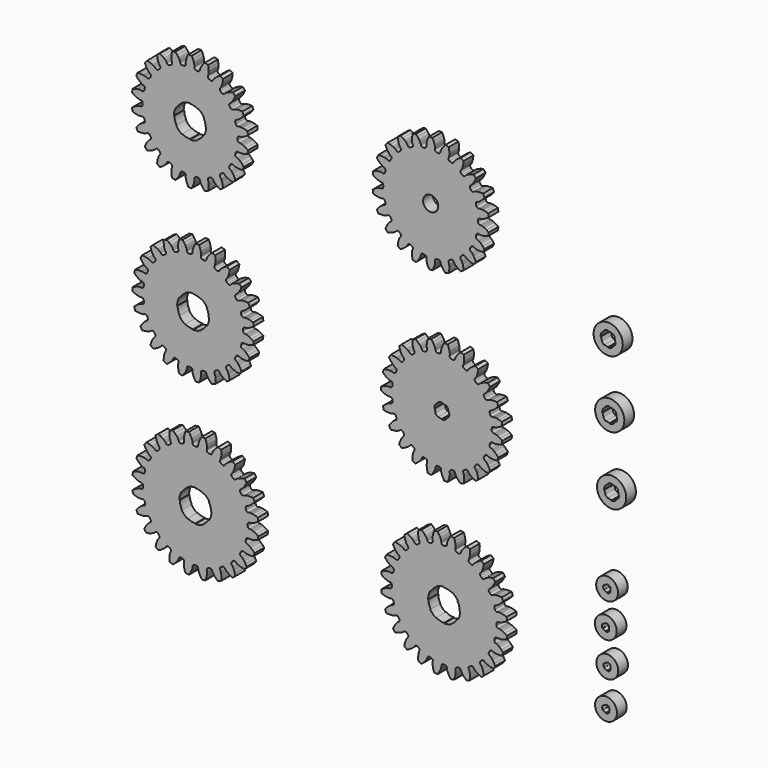
from build123d import *

# Parameters (mm, degrees)
F0_R     = 3.1
F1_DEPTH = 5
F0_R_2   = 6
F0_R_3   = 4.5


# Not quite as in the source:
# - ends of sketch curves that miss each other by under 0.0002 mm in the source are joined


with BuildPart() as f1:
    # F0 (on Front) → F1 (new body)
    with BuildSketch(Plane.XZ):
        with BuildLine():
            ThreePointArc((7.0813803912, 58.2099856207), (7.6127745171, 58.4457380142), (8.1591041791, 58.2470351993))
            ThreePointArc((8.1591041791, 58.2470351993), (8.4227191136, 58.0144167979), (8.6904855572, 57.78658947))
            ThreePointArc((8.6904855572, 57.78658947), (8.9649177305, 57.2740992525), (8.8071907869, 56.7145623918))
            Line((8.8071907869, 56.7145623918), (8.526854, 56.344091))
            Line((8.526854, 56.344091), (8.42499, 56.172609))
            Line((8.42499, 56.172609), (8.304521, 55.931917))
            Line((8.304521, 55.931917), (8.182232, 55.64433))
            Line((8.182232, 55.64433), (8.065432, 55.319895))
            Line((8.065432, 55.319895), (7.95743, 54.963436))
            Line((7.95743, 54.963436), (7.751339, 54.01786))
            Line((7.751339, 54.01786), (7.630041, 52.951038))
            ThreePointArc((7.630041, 52.951038), (8.2171241185, 52.5614483808), (8.8153909693, 52.189259949))
            Line((8.8153909693, 52.189259949), (9.735417, 52.74277))
            Line((9.735417, 52.74277), (10.50993, 53.323043))
            Line((10.50993, 53.323043), (10.789311, 53.569364))
            Line((10.789311, 53.569364), (11.035907, 53.810384))
            Line((11.035907, 53.810384), (11.246705, 54.041091))
            Line((11.246705, 54.041091), (11.415601, 54.25066))
            Line((11.415601, 54.25066), (11.529271, 54.414554))
            Line((11.529271, 54.414554), (11.749807, 54.823457))
            ThreePointArc((11.749807, 54.823457), (12.1932570258, 55.1993709816), (12.7734378249, 55.1626356341))
            ThreePointArc((12.7734378249, 55.1626356341), (13.0919111961, 55.0137091136), (13.4130179103, 54.8705487939))
            ThreePointArc((13.4130179103, 54.8705487939), (13.8207179981, 54.456134629), (13.8270202309, 53.8748269098))
            Line((13.8270202309, 53.8748269098), (13.662412, 53.440381))
            Line((13.662412, 53.440381), (13.612987, 53.247148))
            Line((13.612987, 53.247148), (13.565209, 52.982265))
            Line((13.565209, 52.982265), (13.528895, 52.671874))
            Line((13.528895, 52.671874), (13.50823, 52.327675))
            Line((13.50823, 52.327675), (13.505029, 51.955227))
            Line((13.505029, 51.955227), (13.573686, 50.989891))
            Line((13.573686, 50.989891), (13.75786, 49.93211))
            ThreePointArc((13.75786, 49.93211), (14.4309225964, 49.7237016448), (15.1098129329, 49.535140744))
            Line((15.1098129329, 49.535140744), (15.836629, 50.325431))
            Line((15.836629, 50.325431), (16.416288, 51.100405))
            Line((16.416288, 51.100405), (16.614955, 51.415458))
            Line((16.614955, 51.415458), (16.783659, 51.716189))
            Line((16.783659, 51.716189), (16.92092, 51.99694))
            Line((16.92092, 51.99694), (17.023933, 52.245604))
            Line((17.023933, 52.245604), (17.086823, 52.434883))
            Line((17.086823, 52.434883), (17.183226, 52.889355))
            ThreePointArc((17.183226, 52.889355), (17.5028058412, 53.3749758307), (18.0698338712, 53.5031842062))
            ThreePointArc((18.0698338712, 53.5031842062), (18.4173643789, 53.4500149228), (18.765796976, 53.4031198087))
            ThreePointArc((18.765796976, 53.4031198087), (19.2737371981, 53.1203552676), (19.4435570633, 52.5643689945))
            Line((19.4435570633, 52.5643689945), (19.408014, 52.101147))
            Line((19.408014, 52.101147), (19.415031, 51.901816))
            Line((19.415031, 51.901816), (19.443814, 51.634202))
            Line((19.443814, 51.634202), (19.496419, 51.326153))
            Line((19.496419, 51.326153), (19.573563, 50.990075))
            Line((19.573563, 50.990075), (19.675422, 50.631812))
            Line((19.675422, 50.631812), (20.013265, 49.724922))
            Line((20.013265, 49.724922), (20.48799, 48.761876))
            ThreePointArc((20.48799, 48.761876), (21.192504, 48.751533), (21.8970180104, 48.761875645))
            Line((21.8970180104, 48.761875645), (22.371743, 49.724922))
            Line((22.371743, 49.724922), (22.709586, 50.631812))
            Line((22.709586, 50.631812), (22.811445, 50.990075))
            Line((22.811445, 50.990075), (22.888589, 51.326153))
            Line((22.888589, 51.326153), (22.941194, 51.634202))
            Line((22.941194, 51.634202), (22.969977, 51.901816))
            Line((22.969977, 51.901816), (22.976994, 52.101147))
            Line((22.976994, 52.101147), (22.941452, 52.564369))
            ThreePointArc((22.941452, 52.564369), (23.1112708019, 53.1203552676), (23.619211052, 53.4031205851))
            ThreePointArc((23.619211052, 53.4031205851), (23.9676436211, 53.4500149228), (24.3151741287, 53.5031842067))
            ThreePointArc((24.3151741287, 53.5031842067), (24.8822020776, 53.3749758869), (25.2017821499, 52.8893560302))
            Line((25.2017821499, 52.8893560302), (25.298185, 52.434883))
            Line((25.298185, 52.434883), (25.361075, 52.245604))
            Line((25.361075, 52.245604), (25.464088, 51.99694))
            Line((25.464088, 51.99694), (25.601349, 51.716189))
            Line((25.601349, 51.716189), (25.770053, 51.415458))
            Line((25.770053, 51.415458), (25.96872, 51.100405))
            Line((25.96872, 51.100405), (26.548379, 50.325431))
            Line((26.548379, 50.325431), (27.275195, 49.535141))
            ThreePointArc((27.275195, 49.535141), (27.9540854036, 49.7237016448), (28.6271480164, 49.9321099497))
            Line((28.6271480164, 49.9321099497), (28.811322, 50.989891))
            Line((28.811322, 50.989891), (28.879979, 51.955227))
            Line((28.879979, 51.955227), (28.876778, 52.327675))
            Line((28.876778, 52.327675), (28.856113, 52.671874))
            Line((28.856113, 52.671874), (28.819799, 52.982265))
            Line((28.819799, 52.982265), (28.772021, 53.247148))
            Line((28.772021, 53.247148), (28.722596, 53.440381))
            Line((28.722596, 53.440381), (28.557988, 53.874826))
            ThreePointArc((28.557988, 53.874826), (28.5642900019, 54.456134629), (28.9719901623, 54.8705486269))
            ThreePointArc((28.9719901623, 54.8705486269), (29.2930968039, 55.0137091136), (29.6115703322, 55.1626353059))
            ThreePointArc((29.6115703322, 55.1626353059), (30.1917505461, 55.1993711235), (30.6352009968, 54.8234569983))
            Line((30.6352009968, 54.8234569983), (30.855737, 54.414554))
            Line((30.855737, 54.414554), (30.969407, 54.25066))
            Line((30.969407, 54.25066), (31.138303, 54.041091))
            Line((31.138303, 54.041091), (31.349101, 53.810384))
            Line((31.349101, 53.810384), (31.595697, 53.569364))
            Line((31.595697, 53.569364), (31.875078, 53.323043))
            Line((31.875078, 53.323043), (32.649591, 52.74277))
            Line((32.649591, 52.74277), (33.569617, 52.18926))
            ThreePointArc((33.569617, 52.18926), (34.1678838815, 52.5614483808), (34.7549674089, 52.9510384031))
            Line((34.7549674089, 52.9510384031), (34.633669, 54.01786))
            Line((34.633669, 54.01786), (34.427578, 54.963436))
            Line((34.427578, 54.963436), (34.319576, 55.319895))
            Line((34.319576, 55.319895), (34.202776, 55.64433))
            Line((34.202776, 55.64433), (34.080487, 55.931917))
            Line((34.080487, 55.931917), (33.960018, 56.172609))
            Line((33.960018, 56.172609), (33.858154, 56.344091))
            Line((33.858154, 56.344091), (33.577817, 56.714562))
            ThreePointArc((33.577817, 56.714562), (33.4200903026, 57.2740995564), (33.6945223744, 57.7865895518))
            ThreePointArc((33.6945223744, 57.7865895518), (33.9622888864, 58.0144167979), (34.2259043806, 58.2470345764))
            ThreePointArc((34.2259043806, 58.2470345764), (34.7722331112, 58.4457380269), (35.3036276088, 58.2099856207))
            Line((35.3036276088, 58.2099856207), (35.630432, 57.879778))
            Line((35.630432, 57.879778), (35.785672, 57.754547))
            Line((35.785672, 57.754547), (36.006769, 57.601051))
            Line((36.006769, 57.601051), (36.274026, 57.439078))
            Line((36.274026, 57.439078), (36.578536, 57.277295))
            Line((36.578536, 57.277295), (36.915997, 57.119663))
            Line((36.915997, 57.119663), (37.822618, 56.7811))
            Line((37.822618, 56.7811), (38.861319, 56.509212))
            ThreePointArc((38.861319, 56.509212), (39.3304939405, 57.0348755653), (39.784036163, 57.5740848669))
            Line((39.784036163, 57.5740848669), (39.367093, 58.563519))
            Line((39.367093, 58.563519), (38.902951, 59.41273))
            Line((38.902951, 59.41273), (38.698898, 59.724322))
            Line((38.698898, 59.724322), (38.495425, 60.002709))
            Line((38.495425, 60.002709), (38.297066, 60.244194))
            Line((38.297066, 60.244194), (38.113666, 60.441196))
            Line((38.113666, 60.441196), (37.967617, 60.577033))
            Line((37.967617, 60.577033), (37.594262, 60.853518))
            ThreePointArc((37.594262, 60.853518), (37.2852835326, 61.3459528107), (37.4042140393, 61.9149999737))
            ThreePointArc((37.4042140393, 61.9149999737), (37.5969480529, 62.2090373127), (37.7843494212, 62.5065017399))
            ThreePointArc((37.7843494212, 62.5065017399), (38.2525670658, 62.8510751394), (38.8288550758, 62.7745841339))
            Line((38.8288550758, 62.7745841339), (39.235452, 62.549823))
            Line((39.235452, 62.549823), (39.419685, 62.473401))
            Line((39.419685, 62.473401), (39.675072, 62.388412))
            Line((39.675072, 62.388412), (39.977135, 62.308295))
            Line((39.977135, 62.308295), (40.31489, 62.238856))
            Line((40.31489, 62.238856), (40.683091, 62.182683))
            Line((40.683091, 62.182683), (41.648373, 62.113259))
            Line((41.648373, 62.113259), (42.721598, 62.14502))
            ThreePointArc((42.721598, 62.14502), (43.0236721369, 62.7815732319), (43.3069299749, 63.4267185889))
            Line((43.3069299749, 63.4267185889), (42.62812, 64.258606))
            Line((42.62812, 64.258606), (41.943528, 64.942655))
            Line((41.943528, 64.942655), (41.659955, 65.184137))
            Line((41.659955, 65.184137), (41.386294, 65.393922))
            Line((41.386294, 65.393922), (41.127936, 65.569741))
            Line((41.127936, 65.569741), (40.896463, 65.707094))
            Line((40.896463, 65.707094), (40.71806, 65.796282))
            Line((40.71806, 65.796282), (40.281934, 65.956381))
            ThreePointArc((40.281934, 65.956381), (39.8467359495, 66.3418189833), (39.8005298281, 66.9213227405))
            ThreePointArc((39.8005298281, 66.9213227405), (39.9026170681, 67.2577484229), (39.9986220073, 67.5959607238))
            ThreePointArc((39.9986220073, 67.5959607238), (40.3507965185, 68.0584878061), (40.9252910025, 68.1474540109))
            Line((40.9252910025, 68.1474540109), (41.37874, 68.04635))
            Line((41.37874, 68.04635), (41.577041, 68.024928))
            Line((41.577041, 68.024928), (41.846026, 68.015333))
            Line((41.846026, 68.015333), (42.158426, 68.023562))
            Line((42.158426, 68.023562), (42.502063, 68.052092))
            Line((42.502063, 68.052092), (42.871175, 68.101929))
            Line((42.871175, 68.101929), (43.816914, 68.307269))
            Line((43.816914, 68.307269), (44.837718, 68.640105))
            ThreePointArc((44.837718, 68.640105), (44.9482185585, 69.3359765573), (45.0382440454, 70.0347919948))
            Line((45.0382440454, 70.0347919948), (44.152561, 70.641741))
            Line((44.152561, 70.641741), (43.302981, 71.105208))
            Line((43.302981, 71.105208), (42.962861, 71.257017))
            Line((42.962861, 71.257017), (42.641182, 71.381205))
            Line((42.641182, 71.381205), (42.343755, 71.477114))
            Line((42.343755, 71.477114), (42.082962, 71.54369))
            Line((42.082962, 71.54369), (41.886659, 71.579003))
            Line((41.886659, 71.579003), (41.423093, 71.609746))
            ThreePointArc((41.423093, 71.609746), (40.8969342706, 71.8569618238), (40.6893343545, 72.3999729936))
            ThreePointArc((40.6893343545, 72.3999729936), (40.692504, 72.751533), (40.6893346542, 73.1030930118))
            ThreePointArc((40.6893346542, 73.1030930118), (40.8969342896, 73.6461041968), (41.4230930323, 73.893320425))
            Line((41.4230930323, 73.893320425), (41.886659, 73.924063))
            Line((41.886659, 73.924063), (42.082962, 73.959376))
            Line((42.082962, 73.959376), (42.343755, 74.025952))
            Line((42.343755, 74.025952), (42.641182, 74.121861))
            Line((42.641182, 74.121861), (42.962861, 74.246049))
            Line((42.962861, 74.246049), (43.302981, 74.397858))
            Line((43.302981, 74.397858), (44.152561, 74.861325))
            Line((44.152561, 74.861325), (45.038244, 75.468274))
            ThreePointArc((45.038244, 75.468274), (44.9482184884, 76.1670899303), (44.8377181328, 76.8629620231))
            Line((44.8377181328, 76.8629620231), (43.816914, 77.195797))
            Line((43.816914, 77.195797), (42.871175, 77.401137))
            Line((42.871175, 77.401137), (42.502063, 77.450974))
            Line((42.502063, 77.450974), (42.158426, 77.479504))
            Line((42.158426, 77.479504), (41.846026, 77.487733))
            Line((41.846026, 77.487733), (41.577041, 77.478138))
            Line((41.577041, 77.478138), (41.37874, 77.456716))
            Line((41.37874, 77.456716), (40.925291, 77.355612))
            ThreePointArc((40.925291, 77.355612), (40.3507965185, 77.4445781939), (39.9986219226, 77.9071059788))
            ThreePointArc((39.9986219226, 77.9071059788), (39.9026167978, 78.2453184975), (39.8005299124, 78.5817449725))
            ThreePointArc((39.8005299124, 78.5817449725), (39.8467362373, 79.1612475936), (40.2819333714, 79.5466859556))
            Line((40.2819333714, 79.5466859556), (40.71806, 79.706784))
            Line((40.71806, 79.706784), (40.896463, 79.795972))
            Line((40.896463, 79.795972), (41.127936, 79.933325))
            Line((41.127936, 79.933325), (41.386294, 80.109144))
            Line((41.386294, 80.109144), (41.659955, 80.318929))
            Line((41.659955, 80.318929), (41.943528, 80.560411))
            Line((41.943528, 80.560411), (42.62812, 81.24446))
            Line((42.62812, 81.24446), (43.30693, 82.076348))
            ThreePointArc((43.30693, 82.076348), (43.0236717592, 82.7214935952), (42.7215978789, 83.3580459403))
            Line((42.7215978789, 83.3580459403), (41.648373, 83.389807))
            Line((41.648373, 83.389807), (40.683091, 83.320383))
            Line((40.683091, 83.320383), (40.31489, 83.26421))
            Line((40.31489, 83.26421), (39.977135, 83.194771))
            Line((39.977135, 83.194771), (39.675072, 83.114654))
            Line((39.675072, 83.114654), (39.419685, 83.029665))
            Line((39.419685, 83.029665), (39.235452, 82.953243))
            Line((39.235452, 82.953243), (38.828855, 82.728483))
            ThreePointArc((38.828855, 82.728483), (38.2525668923, 82.6519909051), (37.7843486727, 82.9965647979))
            ThreePointArc((37.7843486727, 82.9965647979), (37.5969475981, 83.2940293948), (37.4042137813, 83.5880668538))
            ThreePointArc((37.4042137813, 83.5880668538), (37.2852835843, 84.1571134781), (37.5942614469, 84.6495483835))
            Line((37.5942614469, 84.6495483835), (37.967617, 84.926033))
            Line((37.967617, 84.926033), (38.113666, 85.06187))
            Line((38.113666, 85.06187), (38.297066, 85.258872))
            Line((38.297066, 85.258872), (38.495425, 85.500357))
            Line((38.495425, 85.500357), (38.698898, 85.778744))
            Line((38.698898, 85.778744), (38.902951, 86.090336))
            Line((38.902951, 86.090336), (39.367093, 86.939547))
            Line((39.367093, 86.939547), (39.784036, 87.928981))
            ThreePointArc((39.784036, 87.928981), (39.3304934458, 88.4681910056), (38.8613183124, 88.9938542872))
            Line((38.8613183124, 88.9938542872), (37.822618, 88.721966))
            Line((37.822618, 88.721966), (36.915997, 88.383403))
            Line((36.915997, 88.383403), (36.578536, 88.225771))
            Line((36.578536, 88.225771), (36.274026, 88.063988))
            Line((36.274026, 88.063988), (36.006769, 87.902015))
            Line((36.006769, 87.902015), (35.785672, 87.748519))
            Line((35.785672, 87.748519), (35.630432, 87.623288))
            Line((35.630432, 87.623288), (35.303628, 87.293081))
            ThreePointArc((35.303628, 87.293081), (34.7722331359, 87.0573279739), (34.2259027705, 87.2560317446))
            ThreePointArc((34.2259027705, 87.2560317446), (33.9622883916, 87.4886496309), (33.6945219508, 87.7164769411))
            ThreePointArc((33.6945219508, 87.7164769411), (33.4200902251, 88.2289671556), (33.577817323, 88.7885037504))
            Line((33.577817323, 88.7885037504), (33.858154, 89.158975))
            Line((33.858154, 89.158975), (33.960018, 89.330457))
            Line((33.960018, 89.330457), (34.080487, 89.571149))
            Line((34.080487, 89.571149), (34.202776, 89.858736))
            Line((34.202776, 89.858736), (34.319576, 90.183171))
            Line((34.319576, 90.183171), (34.427578, 90.53963))
            Line((34.427578, 90.53963), (34.633669, 91.485206))
            Line((34.633669, 91.485206), (34.754967, 92.552028))
            ThreePointArc((34.754967, 92.552028), (34.1678834269, 92.9416179114), (33.5696165889, 93.313806317))
            Line((33.5696165889, 93.313806317), (32.649591, 92.760296))
            Line((32.649591, 92.760296), (31.875078, 92.180023))
            Line((31.875078, 92.180023), (31.595697, 91.933702))
            Line((31.595697, 91.933702), (31.349101, 91.692682))
            Line((31.349101, 91.692682), (31.138303, 91.461975))
            Line((31.138303, 91.461975), (30.969407, 91.252406))
            Line((30.969407, 91.252406), (30.855737, 91.088512))
            Line((30.855737, 91.088512), (30.635201, 90.679609))
            ThreePointArc((30.635201, 90.679609), (30.1917503412, 90.3036948086), (29.6115689721, 90.3404309417))
            ThreePointArc((29.6115689721, 90.3404309417), (29.2930964261, 90.489357059), (28.9719897239, 90.6325173653))
            ThreePointArc((28.9719897239, 90.6325173653), (28.5642897465, 91.0469319853), (28.557988108, 91.6282399578))
            Line((28.557988108, 91.6282399578), (28.722596, 92.062685))
            Line((28.722596, 92.062685), (28.772021, 92.255918))
            Line((28.772021, 92.255918), (28.819799, 92.520801))
            Line((28.819799, 92.520801), (28.856113, 92.831192))
            Line((28.856113, 92.831192), (28.876778, 93.175391))
            Line((28.876778, 93.175391), (28.879979, 93.547839))
            Line((28.879979, 93.547839), (28.811322, 94.513175))
            Line((28.811322, 94.513175), (28.627148, 95.570956))
            ThreePointArc((28.627148, 95.570956), (27.9540851334, 95.7793644345), (27.2751948219, 95.9679253202))
            Line((27.2751948219, 95.9679253202), (26.548379, 95.177635))
            Line((26.548379, 95.177635), (25.96872, 94.402661))
            Line((25.96872, 94.402661), (25.770053, 94.087608))
            Line((25.770053, 94.087608), (25.601349, 93.786877))
            Line((25.601349, 93.786877), (25.464088, 93.506126))
            Line((25.464088, 93.506126), (25.361075, 93.257462))
            Line((25.361075, 93.257462), (25.298185, 93.068183))
            Line((25.298185, 93.068183), (25.201782, 92.613711))
            ThreePointArc((25.201782, 92.613711), (24.8822024147, 92.1280903465), (24.3151739707, 91.9998818195))
            ThreePointArc((24.3151739707, 91.9998818195), (23.9676434803, 92.0530510974), (23.6192109005, 92.0999462067))
            ThreePointArc((23.6192109005, 92.0999462067), (23.1112704497, 92.3827111682), (22.941451023, 92.938697998))
            Line((22.941451023, 92.938697998), (22.976994, 93.401919))
            Line((22.976994, 93.401919), (22.969977, 93.60125))
            Line((22.969977, 93.60125), (22.941194, 93.868864))
            Line((22.941194, 93.868864), (22.888589, 94.176913))
            Line((22.888589, 94.176913), (22.811445, 94.512991))
            Line((22.811445, 94.512991), (22.709586, 94.871254))
            Line((22.709586, 94.871254), (22.371743, 95.778144))
            Line((22.371743, 95.778144), (21.897018, 96.74119))
            ThreePointArc((21.897018, 96.74119), (21.192504, 96.751533), (20.4879900189, 96.7411903558))
            Line((20.4879900189, 96.7411903558), (20.013265, 95.778144))
            Line((20.013265, 95.778144), (19.675422, 94.871254))
            Line((19.675422, 94.871254), (19.573563, 94.512991))
            Line((19.573563, 94.512991), (19.496419, 94.176913))
            Line((19.496419, 94.176913), (19.443814, 93.868864))
            Line((19.443814, 93.868864), (19.415031, 93.60125))
            Line((19.415031, 93.60125), (19.408014, 93.401919))
            Line((19.408014, 93.401919), (19.443556, 92.938697))
            ThreePointArc((19.443556, 92.938697), (19.2737375503, 92.3827111682), (18.7657970714, 92.0999454304))
            ThreePointArc((18.7657970714, 92.0999454304), (18.4173645197, 92.0530510974), (18.0698340294, 91.9998818189))
            ThreePointArc((18.0698340294, 91.9998818189), (17.5028055041, 92.1280904028), (17.1832256174, 92.6137111244))
            Line((17.1832256174, 92.6137111244), (17.086823, 93.068183))
            Line((17.086823, 93.068183), (17.023933, 93.257462))
            Line((17.023933, 93.257462), (16.92092, 93.506126))
            Line((16.92092, 93.506126), (16.783659, 93.786877))
            Line((16.783659, 93.786877), (16.614955, 94.087608))
            Line((16.614955, 94.087608), (16.416288, 94.402661))
            Line((16.416288, 94.402661), (15.836629, 95.177635))
            Line((15.836629, 95.177635), (15.109813, 95.967925))
            ThreePointArc((15.109813, 95.967925), (14.4309228666, 95.7793644345), (13.7578602781, 95.5709561463))
            Line((13.7578602781, 95.5709561463), (13.573686, 94.513175))
            Line((13.573686, 94.513175), (13.505029, 93.547839))
            Line((13.505029, 93.547839), (13.50823, 93.175391))
            Line((13.50823, 93.175391), (13.528895, 92.831192))
            Line((13.528895, 92.831192), (13.565209, 92.520801))
            Line((13.565209, 92.520801), (13.612987, 92.255918))
            Line((13.612987, 92.255918), (13.662412, 92.062685))
            Line((13.662412, 92.062685), (13.82702, 91.62824))
            ThreePointArc((13.82702, 91.62824), (13.8207182535, 91.0469319853), (13.4130182035, 90.6325175322))
            ThreePointArc((13.4130182035, 90.6325175322), (13.0919115739, 90.489357059), (12.7734380572, 90.3404308805))
            ThreePointArc((12.7734380572, 90.3404308805), (12.1932572307, 90.3036949505), (11.7498070032, 90.6796090017))
            Line((11.7498070032, 90.6796090017), (11.529271, 91.088512))
            Line((11.529271, 91.088512), (11.415601, 91.252406))
            Line((11.415601, 91.252406), (11.246705, 91.461975))
            Line((11.246705, 91.461975), (11.035907, 91.692682))
            Line((11.035907, 91.692682), (10.789311, 91.933702))
            Line((10.789311, 91.933702), (10.50993, 92.180023))
            Line((10.50993, 92.180023), (9.735417, 92.760296))
            Line((9.735417, 92.760296), (8.815391, 93.313806))
            ThreePointArc((8.815391, 93.313806), (8.2171245731, 92.9416179114), (7.6300410574, 92.5520279163))
            Line((7.6300410574, 92.5520279163), (7.751339, 91.485206))
            Line((7.751339, 91.485206), (7.95743, 90.53963))
            Line((7.95743, 90.53963), (8.065432, 90.183171))
            Line((8.065432, 90.183171), (8.182232, 89.858736))
            Line((8.182232, 89.858736), (8.304521, 89.571149))
            Line((8.304521, 89.571149), (8.42499, 89.330457))
            Line((8.42499, 89.330457), (8.526854, 89.158975))
            Line((8.526854, 89.158975), (8.807191, 88.788504))
            ThreePointArc((8.807191, 88.788504), (8.964917808, 88.2289674595), (8.6904861176, 87.7164768593))
            ThreePointArc((8.6904861176, 87.7164768593), (8.4227196084, 87.4886496309), (8.1591041166, 87.2560318703))
            ThreePointArc((8.1591041166, 87.2560318703), (7.6127744924, 87.0573279867), (7.0813798914, 87.2930808947))
            Line((7.0813798914, 87.2930808947), (6.754576, 87.623288))
            Line((6.754576, 87.623288), (6.599336, 87.748519))
            Line((6.599336, 87.748519), (6.378239, 87.902015))
            Line((6.378239, 87.902015), (6.110982, 88.063988))
            Line((6.110982, 88.063988), (5.806472, 88.225771))
            Line((5.806472, 88.225771), (5.469011, 88.383403))
            Line((5.469011, 88.383403), (4.56239, 88.721966))
            Line((4.56239, 88.721966), (3.523689, 88.993854))
            ThreePointArc((3.523689, 88.993854), (3.0545143326, 88.4681907498), (2.6009723269, 87.9289817331))
            Line((2.6009723269, 87.9289817331), (3.017915, 86.939547))
            Line((3.017915, 86.939547), (3.482057, 86.090336))
            Line((3.482057, 86.090336), (3.68611, 85.778744))
            Line((3.68611, 85.778744), (3.889583, 85.500357))
            Line((3.889583, 85.500357), (4.087942, 85.258872))
            Line((4.087942, 85.258872), (4.271342, 85.06187))
            Line((4.271342, 85.06187), (4.417391, 84.926033))
            Line((4.417391, 84.926033), (4.790746, 84.649548))
            ThreePointArc((4.790746, 84.649548), (5.0997243444, 84.1571138766), (4.9807939607, 83.5880660263))
            ThreePointArc((4.9807939607, 83.5880660263), (4.7880601096, 83.2940289401), (4.6006587498, 82.996564537))
            ThreePointArc((4.6006587498, 82.996564537), (4.1324406862, 82.6519907969), (3.5561517382, 82.7284825376))
            Line((3.5561517382, 82.7284825376), (3.149556, 82.953243))
            Line((3.149556, 82.953243), (2.965323, 83.029665))
            Line((2.965323, 83.029665), (2.709936, 83.114654))
            Line((2.709936, 83.114654), (2.407873, 83.194771))
            Line((2.407873, 83.194771), (2.070118, 83.26421))
            Line((2.070118, 83.26421), (1.701917, 83.320383))
            Line((1.701917, 83.320383), (0.736635, 83.389807))
            Line((0.736635, 83.389807), (-0.33659, 83.358046))
            ThreePointArc((-0.33659, 83.358046), (-0.6386638399, 82.7214934185), (-0.9219217678, 82.0763479021))
            Line((-0.9219217678, 82.0763479021), (-0.243112, 81.24446))
            Line((-0.243112, 81.24446), (0.44148, 80.560411))
            Line((0.44148, 80.560411), (0.725053, 80.318929))
            Line((0.725053, 80.318929), (0.998714, 80.109144))
            Line((0.998714, 80.109144), (1.257072, 79.933325))
            Line((1.257072, 79.933325), (1.488545, 79.795972))
            Line((1.488545, 79.795972), (1.666948, 79.706784))
            Line((1.666948, 79.706784), (2.103074, 79.546685))
            ThreePointArc((2.103074, 79.546685), (2.5382716191, 79.1612478814), (2.5844783678, 78.5817438848))
            ThreePointArc((2.5844783678, 78.5817438848), (2.4823911228, 78.2453182273), (2.3863861778, 77.9071059513))
            ThreePointArc((2.3863861778, 77.9071059513), (2.0342114815, 77.4445781939), (1.4597169975, 77.3556119891))
            Line((1.4597169975, 77.3556119891), (1.006268, 77.456716))
            Line((1.006268, 77.456716), (0.807967, 77.478138))
            Line((0.807967, 77.478138), (0.538982, 77.487733))
            Line((0.538982, 77.487733), (0.226582, 77.479504))
            Line((0.226582, 77.479504), (-0.117055, 77.450974))
            Line((-0.117055, 77.450974), (-0.486167, 77.401137))
            Line((-0.486167, 77.401137), (-1.431906, 77.195797))
            Line((-1.431906, 77.195797), (-2.45271, 76.862961))
            ThreePointArc((-2.45271, 76.862961), (-2.5632105006, 76.1670898455), (-2.6532360454, 75.4682740052))
            Line((-2.6532360454, 75.4682740052), (-1.767553, 74.861325))
            Line((-1.767553, 74.861325), (-0.917973, 74.397858))
            Line((-0.917973, 74.397858), (-0.577853, 74.246049))
            Line((-0.577853, 74.246049), (-0.256174, 74.121861))
            Line((-0.256174, 74.121861), (0.041253, 74.025952))
            Line((0.041253, 74.025952), (0.302046, 73.959376))
            Line((0.302046, 73.959376), (0.498349, 73.924063))
            Line((0.498349, 73.924063), (0.961915, 73.89332))
            ThreePointArc((0.961915, 73.89332), (1.4880737165, 73.6461041902), (1.6956736452, 73.1030929884))
            ThreePointArc((1.6956736452, 73.1030929884), (1.692504, 72.751533), (1.6956733455, 72.3999730062))
            ThreePointArc((1.6956733455, 72.3999730062), (1.4880737356, 71.8569618304), (0.9619150237, 71.6097455782))
            Line((0.9619150237, 71.6097455782), (0.498349, 71.579003))
            Line((0.498349, 71.579003), (0.302046, 71.54369))
            Line((0.302046, 71.54369), (0.041253, 71.477114))
            Line((0.041253, 71.477114), (-0.256174, 71.381205))
            Line((-0.256174, 71.381205), (-0.577853, 71.257017))
            Line((-0.577853, 71.257017), (-0.917973, 71.105208))
            Line((-0.917973, 71.105208), (-1.767553, 70.641741))
            Line((-1.767553, 70.641741), (-2.653236, 70.034792))
            ThreePointArc((-2.653236, 70.034792), (-2.5632105707, 69.3359766421), (-2.452710331, 68.6401051163))
            Line((-2.452710331, 68.6401051163), (-1.431906, 68.307269))
            Line((-1.431906, 68.307269), (-0.486167, 68.101929))
            Line((-0.486167, 68.101929), (-0.117055, 68.052092))
            Line((-0.117055, 68.052092), (0.226582, 68.023562))
            Line((0.226582, 68.023562), (0.538982, 68.015333))
            Line((0.538982, 68.015333), (0.807967, 68.024928))
            Line((0.807967, 68.024928), (1.006268, 68.04635))
            Line((1.006268, 68.04635), (1.459717, 68.147454))
            ThreePointArc((1.459717, 68.147454), (2.0342114815, 68.0584878061), (2.3863860774, 67.5959600212))
            ThreePointArc((2.3863860774, 67.5959600212), (2.4823908525, 67.2577486932), (2.5844777129, 66.9213222234))
            ThreePointArc((2.5844777129, 66.9213222234), (2.5382719069, 66.3418186955), (2.1030740566, 65.956379841))
            Line((2.1030740566, 65.956379841), (1.666948, 65.796282))
            Line((1.666948, 65.796282), (1.488545, 65.707094))
            Line((1.488545, 65.707094), (1.257072, 65.569741))
            Line((1.257072, 65.569741), (0.998714, 65.393922))
            Line((0.998714, 65.393922), (0.725053, 65.184137))
            Line((0.725053, 65.184137), (0.44148, 64.942655))
            Line((0.44148, 64.942655), (-0.243112, 64.258606))
            Line((-0.243112, 64.258606), (-0.921922, 63.426718))
            ThreePointArc((-0.921922, 63.426718), (-0.6386642176, 62.7815734086), (-0.3365902753, 62.1450208644))
            Line((-0.3365902753, 62.1450208644), (0.736635, 62.113259))
            Line((0.736635, 62.113259), (1.701917, 62.182683))
            Line((1.701917, 62.182683), (2.070118, 62.238856))
            Line((2.070118, 62.238856), (2.407873, 62.308295))
            Line((2.407873, 62.308295), (2.709936, 62.388412))
            Line((2.709936, 62.388412), (2.965323, 62.473401))
            Line((2.965323, 62.473401), (3.149556, 62.549823))
            Line((3.149556, 62.549823), (3.556153, 62.774583))
            ThreePointArc((3.556153, 62.774583), (4.1324405128, 62.8510752476), (4.6006588803, 62.5065019261))
            ThreePointArc((4.6006588803, 62.5065019261), (4.7880596549, 62.2090377675), (4.9807934478, 61.9150002993))
            ThreePointArc((4.9807934478, 61.9150002993), (5.0997243961, 61.3459524122), (4.7907463728, 60.8535174857))
            Line((4.7907463728, 60.8535174857), (4.417391, 60.577033))
            Line((4.417391, 60.577033), (4.271342, 60.441196))
            Line((4.271342, 60.441196), (4.087942, 60.244194))
            Line((4.087942, 60.244194), (3.889583, 60.002709))
            Line((3.889583, 60.002709), (3.68611, 59.724322))
            Line((3.68611, 59.724322), (3.482057, 59.41273))
            Line((3.482057, 59.41273), (3.017915, 58.563519))
            Line((3.017915, 58.563519), (2.600972, 57.574085))
            ThreePointArc((2.600972, 57.574085), (3.0545138379, 57.0348758211), (3.5236887314, 56.5092127531))
            Line((3.5236887314, 56.5092127531), (4.56239, 56.7811))
            Line((4.56239, 56.7811), (5.469011, 57.119663))
            Line((5.469011, 57.119663), (5.806472, 57.277295))
            Line((5.806472, 57.277295), (6.110982, 57.439078))
            Line((6.110982, 57.439078), (6.378239, 57.601051))
            Line((6.378239, 57.601051), (6.599336, 57.754547))
            Line((6.599336, 57.754547), (6.754576, 57.879778))
            Line((6.754576, 57.879778), (7.0813803912, 58.2099856207))
        make_face()
        with Locations((21.192504, 72.751533)):
            Circle(F0_R, mode=Mode.SUBTRACT)
    extrude(amount=F1_DEPTH)


with BuildPart() as f1b:
    # F0 (on Front) → F1, piece 2 (new body)
    with BuildSketch(Plane.XZ):
        with Locations((94.834281, 20.094987)):
            Circle(F0_R_2)
        with BuildLine():
            ThreePointArc((93.2842811075, 22.7796658138), (94.0319420201, 23.0893570776), (94.834281, 23.194987))
            Line((94.834281, 23.194987), (94.834281, 22.994987))
            ThreePointArc((94.834281, 22.994987), (95.5848561513, 22.8961719175), (96.2842808575, 22.6064607532))
            Line((96.2842808575, 22.6064607532), (96.384281, 22.779666))
            ThreePointArc((96.384281, 22.779666), (97.0263118449, 22.2870181985), (97.5189595638, 21.6449873255))
            Line((97.5189595638, 21.6449873255), (97.345754, 21.544987))
            ThreePointArc((97.345754, 21.544987), (97.6354658528, 20.8455623928), (97.734281, 20.094987))
            Line((97.734281, 20.094987), (97.934281, 20.094987))
            ThreePointArc((97.934281, 20.094987), (97.8286510129, 19.2926477787), (97.5189595638, 18.5449866745))
            Line((97.5189595638, 18.5449866745), (97.345754, 18.644987))
            ThreePointArc((97.345754, 18.644987), (96.8848906654, 18.0443773346), (96.2842812905, 17.5835134968))
            Line((96.2842812905, 17.5835134968), (96.384281, 17.410308))
            ThreePointArc((96.384281, 17.410308), (95.6366199799, 17.1006169224), (94.834281, 16.994987))
            Line((94.834281, 16.994987), (94.834281, 17.194987))
            ThreePointArc((94.834281, 17.194987), (94.0837056072, 17.2938021472), (93.3842807095, 17.5835134968))
            Line((93.3842807095, 17.5835134968), (93.284281, 17.410308))
            ThreePointArc((93.284281, 17.410308), (92.6422499783, 17.9029559783), (92.1496021862, 18.5449871075))
            Line((92.1496021862, 18.5449871075), (92.322807, 18.644987))
            ThreePointArc((92.322807, 18.644987), (92.0330960825, 19.3444118487), (91.934281, 20.094987))
            Line((91.934281, 20.094987), (91.734281, 20.094987))
            ThreePointArc((91.734281, 20.094987), (91.8399109224, 20.8973259799), (92.1496021862, 21.6449868925))
            Line((92.1496021862, 21.6449868925), (92.322807, 21.544987))
            ThreePointArc((92.322807, 21.544987), (92.7836713346, 22.1455966654), (93.3842811425, 22.6064607532))
            Line((93.3842811425, 22.6064607532), (93.2842811075, 22.7796658138))
        make_face(mode=Mode.SUBTRACT)
    extrude(amount=F1_DEPTH)


with BuildPart() as f1c:
    # F0 (on Front) → F1, piece 3 (new body)
    with BuildSketch(Plane.XZ):
        with Locations((95.617151, -7.576805)):
            Circle(F0_R_2)
        with BuildLine():
            ThreePointArc((94.0671506745, -4.8921264362), (94.8148117787, -4.5824349871), (95.617151, -4.476805))
            Line((95.617151, -4.476805), (95.617151, -4.676805))
            ThreePointArc((95.617151, -4.676805), (96.3677263928, -4.7756201472), (97.0671512905, -5.0653314968))
            Line((97.0671512905, -5.0653314968), (97.167151, -4.892127))
            ThreePointArc((97.167151, -4.892127), (97.8091821985, -5.3847741551), (98.3018298138, -6.0268051075))
            Line((98.3018298138, -6.0268051075), (98.128625, -6.126805))
            ThreePointArc((98.128625, -6.126805), (98.4183359175, -6.8262298487), (98.517151, -7.576805))
            Line((98.517151, -7.576805), (98.717151, -7.576805))
            ThreePointArc((98.717151, -7.576805), (98.6115210776, -8.3791439799), (98.3018298138, -9.1268048925))
            Line((98.3018298138, -9.1268048925), (98.128625, -9.026805))
            ThreePointArc((98.128625, -9.026805), (97.6677606654, -9.6274146654), (97.0671508575, -10.0882787532))
            Line((97.0671508575, -10.0882787532), (97.167151, -10.261484))
            ThreePointArc((97.167151, -10.261484), (96.4194899799, -10.5711750776), (95.617151, -10.676805))
            Line((95.617151, -10.676805), (95.617151, -10.476805))
            ThreePointArc((95.617151, -10.476805), (94.8665758487, -10.3779899175), (94.1671511425, -10.0882787532))
            Line((94.1671511425, -10.0882787532), (94.067151, -10.261484))
            ThreePointArc((94.067151, -10.261484), (93.4251201551, -9.7688361985), (92.9324724362, -9.1268053255))
            Line((92.9324724362, -9.1268053255), (93.105678, -9.026805))
            ThreePointArc((93.105678, -9.026805), (92.8159661472, -8.3273803928), (92.717151, -7.576805))
            Line((92.717151, -7.576805), (92.517151, -7.576805))
            ThreePointArc((92.517151, -7.576805), (92.6227809871, -6.7744657787), (92.9324724362, -6.0268046745))
            Line((92.9324724362, -6.0268046745), (93.105678, -6.126805))
            ThreePointArc((93.105678, -6.126805), (93.5665413346, -5.5261953346), (94.1671507095, -5.0653314968))
            Line((94.1671507095, -5.0653314968), (94.0671506745, -4.8921264362))
        make_face(mode=Mode.SUBTRACT)
    extrude(amount=F1_DEPTH)


with BuildPart() as f1d:
    # F0 (on Front) → F1, piece 4 (new body)
    with BuildSketch(Plane.XZ):
        with BuildLine():
            ThreePointArc((4.963526029, -75.5581721356), (5.5269996539, -75.6569526548), (5.8638115065, -76.1193571237))
            ThreePointArc((5.8638115065, -76.1193571237), (5.9508828264, -76.4551228115), (6.0433597217, -76.7894400794))
            ThreePointArc((6.0433597217, -76.7894400794), (5.9828742317, -77.3582991681), (5.5442832159, -77.7255826663))
            Line((5.5442832159, -77.7255826663), (5.15385, -77.861651))
            Line((5.15385, -77.861651), (4.893121, -77.991072))
            Line((4.893121, -77.991072), (4.582321, -78.17697))
            Line((4.582321, -78.17697), (4.242597, -78.412037))
            Line((4.242597, -78.412037), (3.885464, -78.691996))
            Line((3.885464, -78.691996), (3.16042, -79.361461))
            Line((3.16042, -79.361461), (2.433315, -80.177067))
            ThreePointArc((2.433315, -80.177067), (2.6974202237, -80.8402824082), (2.9796337297, -81.4959971208))
            Line((2.9796337297, -81.4959971208), (4.070495, -81.558576))
            Line((4.070495, -81.558576), (5.056562, -81.519276))
            Line((5.056562, -81.519276), (5.507054, -81.464705))
            Line((5.507054, -81.464705), (5.913492, -81.390702))
            Line((5.913492, -81.390702), (6.26471, -81.302383))
            Line((6.26471, -81.302383), (6.540589, -81.209534))
            Line((6.540589, -81.209534), (6.912881, -81.029671))
            ThreePointArc((6.912881, -81.029671), (7.4827210244, -80.9792498478), (7.9277345865, -81.3387242299))
            ThreePointArc((7.9277345865, -81.3387242299), (8.0987418275, -81.6405130153), (8.2745952712, -81.9395038375))
            ThreePointArc((8.2745952712, -81.9395038375), (8.3634025295, -82.5046341933), (8.0348162055, -82.9729183171))
            Line((8.0348162055, -82.9729183171), (7.692904, -83.205402))
            Line((7.692904, -83.205402), (7.474555, -83.397896))
            Line((7.474555, -83.397896), (7.22246, -83.6579))
            Line((7.22246, -83.6579), (6.955152, -83.972884))
            Line((6.955152, -83.972884), (6.682646, -84.335737))
            Line((6.682646, -84.335737), (6.155578, -85.170045))
            Line((6.155578, -85.170045), (5.664342, -86.146049))
            ThreePointArc((5.664342, -86.146049), (6.091101003, -86.7183099595), (6.5334100962, -87.2786399219))
            Line((6.5334100962, -87.2786399219), (7.603298, -87.056751))
            Line((7.603298, -87.056751), (8.545593, -86.763577))
            Line((8.545593, -86.763577), (8.966612, -86.59427))
            Line((8.966612, -86.59427), (9.340048, -86.417594))
            Line((9.340048, -86.417594), (9.656439, -86.241383))
            Line((9.656439, -86.241383), (9.898887, -86.080295))
            Line((9.898887, -86.080295), (10.211941, -85.810205))
            ThreePointArc((10.211941, -85.810205), (10.7493135392, -85.6140154126), (11.2722029211, -85.8460630764))
            ThreePointArc((11.2722029211, -85.8460630764), (11.5154917046, -86.0933082956), (11.7627377855, -86.3365972216))
            ThreePointArc((11.7627377855, -86.3365972216), (11.9947855748, -86.8594870898), (11.7985961923, -87.3968591734))
            Line((11.7985961923, -87.3968591734), (11.528506, -87.709914))
            Line((11.528506, -87.709914), (11.367418, -87.952362))
            Line((11.367418, -87.952362), (11.191207, -88.268753))
            Line((11.191207, -88.268753), (11.014531, -88.642189))
            Line((11.014531, -88.642189), (10.845224, -89.063208))
            Line((10.845224, -89.063208), (10.55205, -90.005503))
            Line((10.55205, -90.005503), (10.330161, -91.075391))
            ThreePointArc((10.330161, -91.075391), (10.8904904865, -91.5176995719), (11.4627517598, -91.9444583315))
            Line((11.4627517598, -91.9444583315), (12.438756, -91.453223))
            Line((12.438756, -91.453223), (13.273064, -90.926155))
            Line((13.273064, -90.926155), (13.635917, -90.653649))
            Line((13.635917, -90.653649), (13.950901, -90.386341))
            Line((13.950901, -90.386341), (14.210905, -90.134246))
            Line((14.210905, -90.134246), (14.403399, -89.915897))
            Line((14.403399, -89.915897), (14.635882, -89.573985))
            ThreePointArc((14.635882, -89.573985), (15.1041665418, -89.245398532), (15.6692970962, -89.3342058395))
            ThreePointArc((15.6692970962, -89.3342058395), (15.9682877622, -89.510059044), (16.2700769451, -89.6810660987))
            ThreePointArc((16.2700769451, -89.6810660987), (16.6295511522, -90.1260799756), (16.5791289889, -90.6959189943))
            Line((16.5791289889, -90.6959189943), (16.399267, -91.068212))
            Line((16.399267, -91.068212), (16.306418, -91.344091))
            Line((16.306418, -91.344091), (16.218099, -91.695309))
            Line((16.218099, -91.695309), (16.144096, -92.101747))
            Line((16.144096, -92.101747), (16.089525, -92.552239))
            Line((16.089525, -92.552239), (16.050225, -93.538306))
            Line((16.050225, -93.538306), (16.112804, -94.629167))
            ThreePointArc((16.112804, -94.629167), (16.7685185918, -94.9113807763), (17.4317339918, -95.1754860215))
            Line((17.4317339918, -95.1754860215), (18.24734, -94.448381))
            Line((18.24734, -94.448381), (18.916805, -93.723337))
            Line((18.916805, -93.723337), (19.196764, -93.366204))
            Line((19.196764, -93.366204), (19.431831, -93.02648))
            Line((19.431831, -93.02648), (19.617729, -92.71568))
            Line((19.617729, -92.71568), (19.74715, -92.454951))
            Line((19.74715, -92.454951), (19.883218, -92.064518))
            ThreePointArc((19.883218, -92.064518), (20.2505015749, -91.6259269053), (20.8193607918, -91.5654417297))
            ThreePointArc((20.8193607918, -91.5654417297), (21.1536781885, -91.6579181736), (21.4894438802, -91.744989478))
            ThreePointArc((21.4894438802, -91.744989478), (21.9518480866, -92.0818009311), (22.0506290685, -92.6452740146))
            Line((22.0506290685, -92.6452740146), (21.973252, -93.051433))
            Line((21.973252, -93.051433), (21.954969, -93.341942))
            Line((21.954969, -93.341942), (21.960561, -93.704051))
            Line((21.960561, -93.704051), (21.994274, -94.115794))
            Line((21.994274, -94.115794), (22.058159, -94.56506))
            Line((22.058159, -94.56506), (22.27541, -95.527699))
            Line((22.27541, -95.527699), (22.618193, -96.565194))
            ThreePointArc((22.618193, -96.565194), (23.3246067522, -96.6680793628), (24.0335789327, -96.7515326478))
            Line((24.0335789327, -96.7515326478), (24.633206, -95.838108))
            Line((24.633206, -95.838108), (25.092203, -94.9645))
            Line((25.092203, -94.9645), (25.27019, -94.547077))
            Line((25.27019, -94.547077), (25.409321, -94.158089))
            Line((25.409321, -94.158089), (25.508443, -93.809766))
            Line((25.508443, -93.809766), (25.565973, -93.524423))
            Line((25.565973, -93.524423), (25.596353, -93.112078))
            ThreePointArc((25.596353, -93.112078), (25.8376065895, -92.5933712074), (26.3714279935, -92.3877154034))
            ThreePointArc((26.3714279935, -92.3877154034), (26.718288, -92.390513), (27.0651479979, -92.3877148677))
            ThreePointArc((27.0651479979, -92.3877148677), (27.5989694105, -92.5933712074), (27.8402221222, -93.1120779937))
            Line((27.8402221222, -93.1120779937), (27.870603, -93.524423))
            Line((27.870603, -93.524423), (27.928133, -93.809766))
            Line((27.928133, -93.809766), (28.027255, -94.158089))
            Line((28.027255, -94.158089), (28.166386, -94.547077))
            Line((28.166386, -94.547077), (28.344373, -94.9645))
            Line((28.344373, -94.9645), (28.80337, -95.838108))
            Line((28.80337, -95.838108), (29.402997, -96.751533))
            ThreePointArc((29.402997, -96.751533), (30.1119692478, -96.6680793628), (30.8183830846, -96.5651935296))
            Line((30.8183830846, -96.5651935296), (31.161166, -95.527699))
            Line((31.161166, -95.527699), (31.378417, -94.56506))
            Line((31.378417, -94.56506), (31.442302, -94.115794))
            Line((31.442302, -94.115794), (31.476015, -93.704051))
            Line((31.476015, -93.704051), (31.481607, -93.341942))
            Line((31.481607, -93.341942), (31.463324, -93.051433))
            Line((31.463324, -93.051433), (31.385946, -92.645275))
            ThreePointArc((31.385946, -92.645275), (31.4847279134, -92.0818009311), (31.9471321237, -91.7449894935))
            ThreePointArc((31.9471321237, -91.7449894935), (32.2828978115, -91.6579181736), (32.6172150794, -91.5654412783))
            ThreePointArc((32.6172150794, -91.5654412783), (33.1860744251, -91.6259269053), (33.5533577613, -92.0645180773))
            Line((33.5533577613, -92.0645180773), (33.689426, -92.454951))
            Line((33.689426, -92.454951), (33.818847, -92.71568))
            Line((33.818847, -92.71568), (34.004745, -93.02648))
            Line((34.004745, -93.02648), (34.239812, -93.366204))
            Line((34.239812, -93.366204), (34.519771, -93.723337))
            Line((34.519771, -93.723337), (35.189236, -94.448381))
            Line((35.189236, -94.448381), (36.004842, -95.175486))
            ThreePointArc((36.004842, -95.175486), (36.6680574082, -94.9113807763), (37.3237721208, -94.6291672703))
            Line((37.3237721208, -94.6291672703), (37.386351, -93.538306))
            Line((37.386351, -93.538306), (37.347051, -92.552239))
            Line((37.347051, -92.552239), (37.29248, -92.101747))
            Line((37.29248, -92.101747), (37.218477, -91.695309))
            Line((37.218477, -91.695309), (37.130158, -91.344091))
            Line((37.130158, -91.344091), (37.037309, -91.068212))
            Line((37.037309, -91.068212), (36.857446, -90.69592))
            ThreePointArc((36.857446, -90.69592), (36.8070248478, -90.1260799756), (37.1664992299, -89.6810664135))
            ThreePointArc((37.1664992299, -89.6810664135), (37.4682882378, -89.510059044), (37.7672792784, -89.3342054647))
            ThreePointArc((37.7672792784, -89.3342054647), (38.3324094582, -89.245398532), (38.8006936129, -89.5739852509))
            Line((38.8006936129, -89.5739852509), (39.033177, -89.915897))
            Line((39.033177, -89.915897), (39.225671, -90.134246))
            Line((39.225671, -90.134246), (39.485675, -90.386341))
            Line((39.485675, -90.386341), (39.800659, -90.653649))
            Line((39.800659, -90.653649), (40.163512, -90.926155))
            Line((40.163512, -90.926155), (40.99782, -91.453223))
            Line((40.99782, -91.453223), (41.973824, -91.944459))
            ThreePointArc((41.973824, -91.944459), (42.5460855135, -91.5176995719), (43.1064149219, -91.0753909038))
            Line((43.1064149219, -91.0753909038), (42.884526, -90.005503))
            Line((42.884526, -90.005503), (42.591352, -89.063208))
            Line((42.591352, -89.063208), (42.422045, -88.642189))
            Line((42.422045, -88.642189), (42.245369, -88.268753))
            Line((42.245369, -88.268753), (42.069158, -87.952362))
            Line((42.069158, -87.952362), (41.90807, -87.709914))
            Line((41.90807, -87.709914), (41.63798, -87.39686))
            ThreePointArc((41.63798, -87.39686), (41.4417904252, -86.8594870898), (41.6738380764, -86.3365980789))
            ThreePointArc((41.6738380764, -86.3365980789), (41.9210842954, -86.0933082956), (42.1643732052, -85.8460621987))
            ThreePointArc((42.1643732052, -85.8460621987), (42.6872624608, -85.6140154126), (43.2246347248, -85.8102053051))
            Line((43.2246347248, -85.8102053051), (43.537689, -86.080295))
            Line((43.537689, -86.080295), (43.780137, -86.241383))
            Line((43.780137, -86.241383), (44.096528, -86.417594))
            Line((44.096528, -86.417594), (44.469964, -86.59427))
            Line((44.469964, -86.59427), (44.890983, -86.763577))
            Line((44.890983, -86.763577), (45.833278, -87.056751))
            Line((45.833278, -87.056751), (46.903166, -87.27864))
            ThreePointArc((46.903166, -87.27864), (47.345474997, -86.7183099595), (47.7722341509, -86.1460481094))
            Line((47.7722341509, -86.1460481094), (47.280998, -85.170045))
            Line((47.280998, -85.170045), (46.75393, -84.335737))
            Line((46.75393, -84.335737), (46.481424, -83.972884))
            Line((46.481424, -83.972884), (46.214116, -83.6579))
            Line((46.214116, -83.6579), (45.962021, -83.397896))
            Line((45.962021, -83.397896), (45.743672, -83.205402))
            Line((45.743672, -83.205402), (45.40176, -82.972919))
            ThreePointArc((45.40176, -82.972919), (45.0731734705, -82.5046341933), (45.1619808395, -81.9395039038))
            ThreePointArc((45.1619808395, -81.9395039038), (45.3378341725, -81.6405130153), (45.5088410987, -81.3387240549))
            ThreePointArc((45.5088410987, -81.3387240549), (45.953855208, -80.9792497771), (46.5236939943, -81.0296720111))
            Line((46.5236939943, -81.0296720111), (46.895987, -81.209534))
            Line((46.895987, -81.209534), (47.171866, -81.302383))
            Line((47.171866, -81.302383), (47.523084, -81.390702))
            Line((47.523084, -81.390702), (47.929522, -81.464705))
            Line((47.929522, -81.464705), (48.380014, -81.519276))
            Line((48.380014, -81.519276), (49.366081, -81.558576))
            Line((49.366081, -81.558576), (50.456942, -81.495997))
            ThreePointArc((50.456942, -81.495997), (50.7391557763, -80.8402824082), (51.0032610215, -80.1770670082))
            Line((51.0032610215, -80.1770670082), (50.276156, -79.361461))
            Line((50.276156, -79.361461), (49.551112, -78.691996))
            Line((49.551112, -78.691996), (49.193979, -78.412037))
            Line((49.193979, -78.412037), (48.854255, -78.17697))
            Line((48.854255, -78.17697), (48.543455, -77.991072))
            Line((48.543455, -77.991072), (48.282726, -77.861651))
            Line((48.282726, -77.861651), (47.892293, -77.725583))
            ThreePointArc((47.892293, -77.725583), (47.4537017683, -77.3582991681), (47.393216805, -76.7894399444))
            ThreePointArc((47.393216805, -76.7894399444), (47.4856932051, -76.4551226941), (47.5727645371, -76.1193568839))
            ThreePointArc((47.5727645371, -76.1193568839), (47.9095764493, -75.6569525905), (48.473049971, -75.5581721356))
            Line((48.473049971, -75.5581721356), (48.879208, -75.635549))
            Line((48.879208, -75.635549), (49.169717, -75.653832))
            Line((49.169717, -75.653832), (49.531826, -75.64824))
            Line((49.531826, -75.64824), (49.943569, -75.614527))
            Line((49.943569, -75.614527), (50.392835, -75.550642))
            Line((50.392835, -75.550642), (51.355474, -75.333391))
            Line((51.355474, -75.333391), (52.392969, -74.990608))
            ThreePointArc((52.392969, -74.990608), (52.4958543798, -74.2841941184), (52.5793076585, -73.5752219645))
            Line((52.5793076585, -73.5752219645), (51.665883, -72.975595))
            Line((51.665883, -72.975595), (50.792275, -72.516598))
            Line((50.792275, -72.516598), (50.374852, -72.338611))
            Line((50.374852, -72.338611), (49.985864, -72.19948))
            Line((49.985864, -72.19948), (49.637541, -72.100358))
            Line((49.637541, -72.100358), (49.352198, -72.042828))
            Line((49.352198, -72.042828), (48.939853, -72.012448))
            ThreePointArc((48.939853, -72.012448), (48.4211462074, -71.7711944105), (48.2154904034, -71.2373730065))
            ThreePointArc((48.2154904034, -71.2373730065), (48.218288, -70.890513), (48.2154898677, -70.5436530021))
            ThreePointArc((48.2154898677, -70.5436530021), (48.4211462074, -70.0098315895), (48.9398529937, -69.7685788778))
            Line((48.9398529937, -69.7685788778), (49.352198, -69.738198))
            Line((49.352198, -69.738198), (49.637541, -69.680668))
            Line((49.637541, -69.680668), (49.985864, -69.581546))
            Line((49.985864, -69.581546), (50.374852, -69.442415))
            Line((50.374852, -69.442415), (50.792275, -69.264428))
            Line((50.792275, -69.264428), (51.665883, -68.805431))
            Line((51.665883, -68.805431), (52.579308, -68.205804))
            ThreePointArc((52.579308, -68.205804), (52.4958543798, -67.4968318816), (52.3929685545, -66.7904180711))
            Line((52.3929685545, -66.7904180711), (51.355474, -66.447635))
            Line((51.355474, -66.447635), (50.392835, -66.230384))
            Line((50.392835, -66.230384), (49.943569, -66.166499))
            Line((49.943569, -66.166499), (49.531826, -66.132786))
            Line((49.531826, -66.132786), (49.169717, -66.127194))
            Line((49.169717, -66.127194), (48.879208, -66.145477))
            Line((48.879208, -66.145477), (48.47305, -66.222855))
            ThreePointArc((48.47305, -66.222855), (47.9095764493, -66.1240734095), (47.5727645527, -65.6616691122))
            ThreePointArc((47.5727645527, -65.6616691122), (47.4856932051, -65.3259033059), (47.3932162783, -64.9915859206))
            ThreePointArc((47.3932162783, -64.9915859206), (47.4537018408, -64.4227266959), (47.8922930773, -64.0554432387))
            Line((47.8922930773, -64.0554432387), (48.282726, -63.919375))
            Line((48.282726, -63.919375), (48.543455, -63.789954))
            Line((48.543455, -63.789954), (48.854255, -63.604056))
            Line((48.854255, -63.604056), (49.193979, -63.368989))
            Line((49.193979, -63.368989), (49.551112, -63.08903))
            Line((49.551112, -63.08903), (50.276156, -62.419565))
            Line((50.276156, -62.419565), (51.003261, -61.603959))
            ThreePointArc((51.003261, -61.603959), (50.7391557763, -60.9407435918), (50.4569422703, -60.2850288792))
            Line((50.4569422703, -60.2850288792), (49.366081, -60.22245))
            Line((49.366081, -60.22245), (48.380014, -60.26175))
            Line((48.380014, -60.26175), (47.929522, -60.316321))
            Line((47.929522, -60.316321), (47.523084, -60.390324))
            Line((47.523084, -60.390324), (47.171866, -60.478643))
            Line((47.171866, -60.478643), (46.895987, -60.571492))
            Line((46.895987, -60.571492), (46.523695, -60.751355))
            ThreePointArc((46.523695, -60.751355), (45.9538550075, -60.8017761619), (45.508841225, -60.442301431))
            ThreePointArc((45.508841225, -60.442301431), (45.3378341725, -60.1405129847), (45.1619807288, -59.8415221625))
            ThreePointArc((45.1619807288, -59.8415221625), (45.073173532, -59.2763915418), (45.4017602509, -58.8081073871))
            Line((45.4017602509, -58.8081073871), (45.743672, -58.575624))
            Line((45.743672, -58.575624), (45.962021, -58.38313))
            Line((45.962021, -58.38313), (46.214116, -58.123126))
            Line((46.214116, -58.123126), (46.481424, -57.808142))
            Line((46.481424, -57.808142), (46.75393, -57.445289))
            Line((46.75393, -57.445289), (47.280998, -56.610981))
            Line((47.280998, -56.610981), (47.772234, -55.634977))
            ThreePointArc((47.772234, -55.634977), (47.3454747505, -55.0627157193), (46.9031659038, -54.5023860781))
            Line((46.9031659038, -54.5023860781), (45.833278, -54.724275))
            Line((45.833278, -54.724275), (44.890983, -55.017449))
            Line((44.890983, -55.017449), (44.469964, -55.186756))
            Line((44.469964, -55.186756), (44.096528, -55.363432))
            Line((44.096528, -55.363432), (43.780137, -55.539643))
            Line((43.780137, -55.539643), (43.537689, -55.700731))
            Line((43.537689, -55.700731), (43.224635, -55.970821))
            ThreePointArc((43.224635, -55.970821), (42.6872627955, -56.1670105987), (42.1643730789, -55.9349629236))
            ThreePointArc((42.1643730789, -55.9349629236), (41.9210837955, -55.6877172045), (41.6738377148, -55.4444282945))
            ThreePointArc((41.6738377148, -55.4444282945), (41.4417904126, -54.9215385392), (41.6379803051, -54.3841662752))
            Line((41.6379803051, -54.3841662752), (41.90807, -54.071112))
            Line((41.90807, -54.071112), (42.069158, -53.828664))
            Line((42.069158, -53.828664), (42.245369, -53.512273))
            Line((42.245369, -53.512273), (42.422045, -53.138837))
            Line((42.422045, -53.138837), (42.591352, -52.717818))
            Line((42.591352, -52.717818), (42.884526, -51.775523))
            Line((42.884526, -51.775523), (43.106415, -50.705635))
            ThreePointArc((43.106415, -50.705635), (42.5460852807, -50.2633262495), (41.9738237651, -49.8365673242))
            Line((41.9738237651, -49.8365673242), (40.99782, -50.327803))
            Line((40.99782, -50.327803), (40.163512, -50.854871))
            Line((40.163512, -50.854871), (39.800659, -51.127377))
            Line((39.800659, -51.127377), (39.485675, -51.394685))
            Line((39.485675, -51.394685), (39.225671, -51.64678))
            Line((39.225671, -51.64678), (39.033177, -51.865129))
            Line((39.033177, -51.865129), (38.800694, -52.207041))
            ThreePointArc((38.800694, -52.207041), (38.3324098669, -52.5356273732), (37.7672789038, -52.4468201605))
            ThreePointArc((37.7672789038, -52.4468201605), (37.4682880153, -52.2709668275), (37.1664990549, -52.0999599013))
            ThreePointArc((37.1664990549, -52.0999599013), (36.8070246473, -51.654945366), (36.8574474161, -51.0851062125))
            Line((36.8574474161, -51.0851062125), (37.037309, -50.712814))
            Line((37.037309, -50.712814), (37.130158, -50.436935))
            Line((37.130158, -50.436935), (37.218477, -50.085717))
            Line((37.218477, -50.085717), (37.29248, -49.679279))
            Line((37.29248, -49.679279), (37.347051, -49.228787))
            Line((37.347051, -49.228787), (37.386351, -48.24272))
            Line((37.386351, -48.24272), (37.323772, -47.151859))
            ThreePointArc((37.323772, -47.151859), (36.6680572197, -46.8696451457), (36.0048420082, -46.6055399785))
            Line((36.0048420082, -46.6055399785), (35.189236, -47.332645))
            Line((35.189236, -47.332645), (34.519771, -48.057689))
            Line((34.519771, -48.057689), (34.239812, -48.414822))
            Line((34.239812, -48.414822), (34.004745, -48.754546))
            Line((34.004745, -48.754546), (33.818847, -49.065346))
            Line((33.818847, -49.065346), (33.689426, -49.326075))
            Line((33.689426, -49.326075), (33.553358, -49.716508))
            ThreePointArc((33.553358, -49.716508), (33.1860743041, -50.1550991592), (32.6172149444, -50.215584195))
            ThreePointArc((32.6172149444, -50.215584195), (32.2828975616, -50.1231077594), (31.9471318839, -50.0360364629))
            ThreePointArc((31.9471318839, -50.0360364629), (31.4847275905, -49.6992245507), (31.3859471356, -49.135751029))
            Line((31.3859471356, -49.135751029), (31.463324, -48.729593))
            Line((31.463324, -48.729593), (31.481607, -48.439084))
            Line((31.481607, -48.439084), (31.476015, -48.076975))
            Line((31.476015, -48.076975), (31.442302, -47.665232))
            Line((31.442302, -47.665232), (31.378417, -47.215966))
            Line((31.378417, -47.215966), (31.161166, -46.253327))
            Line((31.161166, -46.253327), (30.818383, -45.215832))
            ThreePointArc((30.818383, -45.215832), (30.1119691184, -45.1129466202), (29.4029969645, -45.0294933415))
            Line((29.4029969645, -45.0294933415), (28.80337, -45.942918))
            Line((28.80337, -45.942918), (28.344373, -46.816526))
            Line((28.344373, -46.816526), (28.166386, -47.233949))
            Line((28.166386, -47.233949), (28.027255, -47.622937))
            Line((28.027255, -47.622937), (27.928133, -47.97126))
            Line((27.928133, -47.97126), (27.870603, -48.256603))
            Line((27.870603, -48.256603), (27.840223, -48.668948))
            ThreePointArc((27.840223, -48.668948), (27.5989694046, -49.1876547981), (27.0651479904, -49.3933105964))
            ThreePointArc((27.0651479904, -49.3933105964), (26.718288, -49.390513), (26.3714280021, -49.3933111323))
            ThreePointArc((26.3714280021, -49.3933111323), (25.8376065954, -49.1876547981), (25.5963538778, -48.6689480063))
            Line((25.5963538778, -48.6689480063), (25.565973, -48.256603))
            Line((25.565973, -48.256603), (25.508443, -47.97126))
            Line((25.508443, -47.97126), (25.409321, -47.622937))
            Line((25.409321, -47.622937), (25.27019, -47.233949))
            Line((25.27019, -47.233949), (25.092203, -46.816526))
            Line((25.092203, -46.816526), (24.633206, -45.942918))
            Line((24.633206, -45.942918), (24.033579, -45.029493))
            ThreePointArc((24.033579, -45.029493), (23.3246068816, -45.1129466202), (22.6181930711, -45.2158324455))
            Line((22.6181930711, -45.2158324455), (22.27541, -46.253327))
            Line((22.27541, -46.253327), (22.058159, -47.215966))
            Line((22.058159, -47.215966), (21.994274, -47.665232))
            Line((21.994274, -47.665232), (21.960561, -48.076975))
            Line((21.960561, -48.076975), (21.954969, -48.439084))
            Line((21.954969, -48.439084), (21.973252, -48.729593))
            Line((21.973252, -48.729593), (22.05063, -49.135751))
            ThreePointArc((22.05063, -49.135751), (21.9518484095, -49.6992245507), (21.4894441122, -50.0360364473))
            ThreePointArc((21.4894441122, -50.0360364473), (21.1536784384, -50.1231077594), (20.8193611844, -50.2155846464))
            ThreePointArc((20.8193611844, -50.2155846464), (20.2505016959, -50.1550991592), (19.8832182387, -49.7165079227))
            Line((19.8832182387, -49.7165079227), (19.74715, -49.326075))
            Line((19.74715, -49.326075), (19.617729, -49.065346))
            Line((19.617729, -49.065346), (19.431831, -48.754546))
            Line((19.431831, -48.754546), (19.196764, -48.414822))
            Line((19.196764, -48.414822), (18.916805, -48.057689))
            Line((18.916805, -48.057689), (18.24734, -47.332645))
            Line((18.24734, -47.332645), (17.431734, -46.60554))
            ThreePointArc((17.431734, -46.60554), (16.7685187803, -46.8696451457), (16.1128042517, -47.1518585633))
            Line((16.1128042517, -47.1518585633), (16.050225, -48.24272))
            Line((16.050225, -48.24272), (16.089525, -49.228787))
            Line((16.089525, -49.228787), (16.144096, -49.679279))
            Line((16.144096, -49.679279), (16.218099, -50.085717))
            Line((16.218099, -50.085717), (16.306418, -50.436935))
            Line((16.306418, -50.436935), (16.399267, -50.712814))
            Line((16.399267, -50.712814), (16.57913, -51.085106))
            ThreePointArc((16.57913, -51.085106), (16.6295513527, -51.654945366), (16.2700771948, -52.0999593503))
            ThreePointArc((16.2700771948, -52.0999593503), (15.9682879847, -52.2709668275), (15.6692971625, -52.4468202712))
            ThreePointArc((15.6692971625, -52.4468202712), (15.1041661331, -52.5356273732), (14.6358819307, -52.2070400449))
            Line((14.6358819307, -52.2070400449), (14.403399, -51.865129))
            Line((14.403399, -51.865129), (14.210905, -51.64678))
            Line((14.210905, -51.64678), (13.950901, -51.394685))
            Line((13.950901, -51.394685), (13.635917, -51.127377))
            Line((13.635917, -51.127377), (13.273064, -50.854871))
            Line((13.273064, -50.854871), (12.438756, -50.327803))
            Line((12.438756, -50.327803), (11.462752, -49.836567))
            ThreePointArc((11.462752, -49.836567), (10.8904907193, -50.2633262495), (10.3301610781, -50.7056350962))
            Line((10.3301610781, -50.7056350962), (10.55205, -51.775523))
            Line((10.55205, -51.775523), (10.845224, -52.717818))
            Line((10.845224, -52.717818), (11.014531, -53.138837))
            Line((11.014531, -53.138837), (11.191207, -53.512273))
            Line((11.191207, -53.512273), (11.367418, -53.828664))
            Line((11.367418, -53.828664), (11.528506, -54.071112))
            Line((11.528506, -54.071112), (11.798596, -54.384166))
            ThreePointArc((11.798596, -54.384166), (11.9947855874, -54.9215385392), (11.7627379236, -55.4444279211))
            ThreePointArc((11.7627379236, -55.4444279211), (11.5154922045, -55.6877172045), (11.2722032945, -55.9349632852))
            ThreePointArc((11.2722032945, -55.9349632852), (10.7493132045, -56.1670105987), (10.2119407778, -55.9708202463))
            Line((10.2119407778, -55.9708202463), (9.898887, -55.700731))
            Line((9.898887, -55.700731), (9.656439, -55.539643))
            Line((9.656439, -55.539643), (9.340048, -55.363432))
            Line((9.340048, -55.363432), (8.966612, -55.186756))
            Line((8.966612, -55.186756), (8.545593, -55.017449))
            Line((8.545593, -55.017449), (7.603298, -54.724275))
            Line((7.603298, -54.724275), (6.53341, -54.502386))
            ThreePointArc((6.53341, -54.502386), (6.0911012495, -55.0627157193), (5.6643423242, -55.6349772349))
            Line((5.6643423242, -55.6349772349), (6.155578, -56.610981))
            Line((6.155578, -56.610981), (6.682646, -57.445289))
            Line((6.682646, -57.445289), (6.955152, -57.808142))
            Line((6.955152, -57.808142), (7.22246, -58.123126))
            Line((7.22246, -58.123126), (7.474555, -58.38313))
            Line((7.474555, -58.38313), (7.692904, -58.575624))
            Line((7.692904, -58.575624), (8.034816, -58.808107))
            ThreePointArc((8.034816, -58.808107), (8.363402468, -59.2763915418), (8.2745951605, -59.8415220962))
            ThreePointArc((8.2745951605, -59.8415220962), (8.0987418275, -60.1405129847), (7.9277349013, -60.4423019451))
            ThreePointArc((7.9277349013, -60.4423019451), (7.4827212249, -60.8017760911), (6.9128816006, -60.7513537821))
            Line((6.9128816006, -60.7513537821), (6.540589, -60.571492))
            Line((6.540589, -60.571492), (6.26471, -60.478643))
            Line((6.26471, -60.478643), (5.913492, -60.390324))
            Line((5.913492, -60.390324), (5.507054, -60.316321))
            Line((5.507054, -60.316321), (5.056562, -60.26175))
            Line((5.056562, -60.26175), (4.070495, -60.22245))
            Line((4.070495, -60.22245), (2.979634, -60.285029))
            ThreePointArc((2.979634, -60.285029), (2.6974202237, -60.9407435918), (2.4333149785, -61.6039589918))
            Line((2.4333149785, -61.6039589918), (3.16042, -62.419565))
            Line((3.16042, -62.419565), (3.885464, -63.08903))
            Line((3.885464, -63.08903), (4.242597, -63.368989))
            Line((4.242597, -63.368989), (4.582321, -63.604056))
            Line((4.582321, -63.604056), (4.893121, -63.789954))
            Line((4.893121, -63.789954), (5.15385, -63.919375))
            Line((5.15385, -63.919375), (5.544283, -64.055443))
            ThreePointArc((5.544283, -64.055443), (5.9828741592, -64.4227266959), (6.043359195, -64.9915860556))
            ThreePointArc((6.043359195, -64.9915860556), (5.9508828264, -65.3259031885), (5.863811522, -65.6616688802))
            ThreePointArc((5.863811522, -65.6616688802), (5.5269996539, -66.1240733452), (4.963526029, -66.2228538644))
            Line((4.963526029, -66.2228538644), (4.557368, -66.145477))
            Line((4.557368, -66.145477), (4.266859, -66.127194))
            Line((4.266859, -66.127194), (3.90475, -66.132786))
            Line((3.90475, -66.132786), (3.493007, -66.166499))
            Line((3.493007, -66.166499), (3.043741, -66.230384))
            Line((3.043741, -66.230384), (2.081102, -66.447635))
            Line((2.081102, -66.447635), (1.043607, -66.790418))
            ThreePointArc((1.043607, -66.790418), (0.9407216305, -67.4968318034), (0.8572683415, -68.2058040355))
            Line((0.8572683415, -68.2058040355), (1.770693, -68.805431))
            Line((1.770693, -68.805431), (2.644301, -69.264428))
            Line((2.644301, -69.264428), (3.061724, -69.442415))
            Line((3.061724, -69.442415), (3.450712, -69.581546))
            Line((3.450712, -69.581546), (3.799035, -69.680668))
            Line((3.799035, -69.680668), (4.084378, -69.738198))
            Line((4.084378, -69.738198), (4.496723, -69.768578))
            ThreePointArc((4.496723, -69.768578), (5.0154297926, -70.0098315895), (5.2210855966, -70.5436529935))
            ThreePointArc((5.2210855966, -70.5436529935), (5.218288, -70.890513), (5.2210861323, -71.2373729979))
            ThreePointArc((5.2210861323, -71.2373729979), (5.0154297926, -71.7711944105), (4.4967230063, -72.0124471222))
            Line((4.4967230063, -72.0124471222), (4.084378, -72.042828))
            Line((4.084378, -72.042828), (3.799035, -72.100358))
            Line((3.799035, -72.100358), (3.450712, -72.19948))
            Line((3.450712, -72.19948), (3.061724, -72.338611))
            Line((3.061724, -72.338611), (2.644301, -72.516598))
            Line((2.644301, -72.516598), (1.770693, -72.975595))
            Line((1.770693, -72.975595), (0.857268, -73.575222))
            ThreePointArc((0.857268, -73.575222), (0.9407216305, -74.2841941966), (1.0436074704, -74.9906080846))
            Line((1.0436074704, -74.9906080846), (2.081102, -75.333391))
            Line((2.081102, -75.333391), (3.043741, -75.550642))
            Line((3.043741, -75.550642), (3.493007, -75.614527))
            Line((3.493007, -75.614527), (3.90475, -75.64824))
            Line((3.90475, -75.64824), (4.266859, -75.653832))
            Line((4.266859, -75.653832), (4.557368, -75.635549))
            Line((4.557368, -75.635549), (4.963526029, -75.5581721356))
        make_face()
        with BuildLine():
            ThreePointArc((23.4182881451, -65.1747452513), (25.0100823832, -64.5154025248), (26.718288, -64.290513))
            Line((26.718288, -64.290513), (26.718288, -64.490513))
            ThreePointArc((26.718288, -64.490513), (28.3747297883, -64.7085876848), (29.91828782, -65.3479503118))
            Line((29.91828782, -65.3479503118), (30.018288, -65.174745))
            ThreePointArc((30.018288, -65.174745), (31.3851927558, -66.2236082442), (32.4340557487, -67.5905131451))
            Line((32.4340557487, -67.5905131451), (32.260851, -67.690513))
            ThreePointArc((32.260851, -67.690513), (32.9002133152, -69.2340712117), (33.118288, -70.890513))
            Line((33.118288, -70.890513), (33.318288, -70.890513))
            ThreePointArc((33.318288, -70.890513), (33.0933984752, -72.5987186168), (32.4340557487, -74.1905128549))
            Line((32.4340557487, -74.1905128549), (32.260851, -74.090513))
            ThreePointArc((32.260851, -74.090513), (31.2437715764, -75.4159962228), (29.918288253, -76.4330754382))
            Line((29.918288253, -76.4330754382), (30.018288, -76.60628))
            ThreePointArc((30.018288, -76.60628), (28.4264938583, -77.2656234105), (26.718288, -77.490513))
            Line((26.718288, -77.490513), (26.718288, -77.290513))
            ThreePointArc((26.718288, -77.290513), (25.0618459703, -77.0724382504), (23.518287747, -76.4330754382))
            Line((23.518287747, -76.4330754382), (23.418288, -76.60628))
            ThreePointArc((23.418288, -76.60628), (22.0513830674, -75.5574175791), (21.0025202513, -74.1905128549))
            Line((21.0025202513, -74.1905128549), (21.175726, -74.090513))
            ThreePointArc((21.175726, -74.090513), (20.5363627496, -72.5469550297), (20.318288, -70.890513))
            Line((20.318288, -70.890513), (20.118288, -70.890513))
            ThreePointArc((20.118288, -70.890513), (20.3431775248, -69.1823073832), (21.0025202513, -67.5905131451))
            Line((21.0025202513, -67.5905131451), (21.175726, -67.690513))
            ThreePointArc((21.175726, -67.690513), (22.1928047772, -66.3650294236), (23.51828818, -65.3479503118))
            Line((23.51828818, -65.3479503118), (23.4182881451, -65.1747452513))
        make_face(mode=Mode.SUBTRACT)
    extrude(amount=F1_DEPTH)


with BuildPart() as f1e:
    # F0 (on Front) → F1, piece 5 (new body)
    with BuildSketch(Plane.XZ):
        with BuildLine():
            ThreePointArc((8.6115728195, -13.4079537521), (9.1709588577, -13.2675897833), (9.6710783171, -13.5548097509))
            ThreePointArc((9.6710783171, -13.5548097509), (9.8893314127, -13.8277997015), (10.1122063659, -14.0970286918))
            ThreePointArc((10.1122063659, -14.0970286918), (10.2916672152, -14.6451245394), (10.0404291436, -15.1642531584))
            Line((10.0404291436, -15.1642531584), (9.730002, -15.452773))
            Line((9.730002, -15.452773), (9.595535, -15.609589))
            Line((9.595535, -15.609589), (9.431849, -15.829619))
            Line((9.431849, -15.829619), (9.258147, -16.094994))
            Line((9.258147, -16.094994), (9.083285, -16.397223))
            Line((9.083285, -16.397223), (8.911206, -16.73231))
            Line((8.911206, -16.73231), (8.533576, -17.633959))
            Line((8.533576, -17.633959), (8.216223, -18.670056))
            ThreePointArc((8.216223, -18.670056), (8.7275844731, -19.161396157), (9.2526760346, -19.6380349608))
            Line((9.2526760346, -19.6380349608), (10.2647, -19.250717))
            Line((10.2647, -19.250717), (11.138477, -18.812435))
            Line((11.138477, -18.812435), (11.46104, -18.617891))
            Line((11.46104, -18.617891), (11.750632, -18.422812))
            Line((11.750632, -18.422812), (12.003534, -18.231405))
            Line((12.003534, -18.231405), (12.211881, -18.053085))
            Line((12.211881, -18.053085), (12.359155, -17.90823))
            Line((12.359155, -17.90823), (12.625817, -17.578837))
            ThreePointArc((12.625817, -17.578837), (13.1265902924, -17.2927586057), (13.6856552524, -17.4343976551))
            ThreePointArc((13.6856552524, -17.4343976551), (13.969466495, -17.6383798762), (14.25671384, -17.8374942351))
            ThreePointArc((14.25671384, -17.8374942351), (14.5773934283, -18.31684729), (14.4755311673, -18.8845081052))
            Line((14.4755311673, -18.8845081052), (14.254458, -19.246081))
            Line((14.254458, -19.246081), (14.167286, -19.43336))
            Line((14.167286, -19.43336), (14.069032, -19.689393))
            Line((14.069032, -19.689393), (13.973369, -19.991791))
            Line((13.973369, -19.991791), (13.886532, -20.32999))
            Line((13.886532, -20.32999), (13.81124, -20.699078))
            Line((13.81124, -20.699078), (13.690875, -21.669175))
            Line((13.690875, -21.669175), (13.664827, -22.752471))
            ThreePointArc((13.664827, -22.752471), (14.2897870964, -23.0876274806), (14.9240019996, -23.4049230009))
            Line((14.9240019996, -23.4049230009), (15.794001, -22.758927))
            Line((15.794001, -22.758927), (16.517129, -22.101156))
            Line((16.517129, -22.101156), (16.775243, -21.8268))
            Line((16.775243, -21.8268), (17.001464, -21.560824))
            Line((17.001464, -21.560824), (17.193347, -21.308283))
            Line((17.193347, -21.308283), (17.345857, -21.080363))
            Line((17.345857, -21.080363), (17.448589, -20.901146))
            Line((17.448589, -20.901146), (17.616494, -20.512024))
            ThreePointArc((17.616494, -20.512024), (18.0215136778, -20.1014461729), (18.5980611799, -20.0869995199))
            ThreePointArc((18.5980611799, -20.0869995199), (18.9263812173, -20.2068459983), (19.2566969316, -20.3210782035))
            ThreePointArc((19.2566969316, -20.3210782035), (19.6948131849, -20.6961371962), (19.749880518, -21.2702301534))
            Line((19.749880518, -21.2702301534), (19.634557, -21.678039))
            Line((19.634557, -21.678039), (19.601145, -21.881893))
            Line((19.601145, -21.881893), (19.575611, -22.154939))
            Line((19.575611, -22.154939), (19.565082, -22.471934))
            Line((19.565082, -22.471934), (19.57271, -22.82102))
            Line((19.57271, -22.82102), (19.599789, -23.196734))
            Line((19.599789, -23.196734), (19.745616, -24.163331))
            Line((19.745616, -24.163331), (20.012803, -25.213483))
            ThreePointArc((20.012803, -25.213483), (20.7050127291, -25.3675992036), (21.4013150872, -25.5020195111))
            Line((21.4013150872, -25.5020195111), (22.064764, -24.645256))
            Line((22.064764, -24.645256), (22.583612, -23.816779))
            Line((22.583612, -23.816779), (22.758134, -23.482958))
            Line((22.758134, -23.482958), (22.904206, -23.165812))
            Line((22.904206, -23.165812), (23.020839, -22.870866))
            Line((23.020839, -22.870866), (23.106202, -22.610252))
            Line((23.106202, -22.610252), (23.156772, -22.409964))
            Line((23.156772, -22.409964), (23.213466, -21.989971))
            ThreePointArc((23.213466, -21.989971), (23.4926945667, -21.485345412), (24.043964044, -21.3158834862))
            ThreePointArc((24.043964044, -21.3158834862), (24.3924436917, -21.3427067797), (24.7413300082, -21.3635848401))
            ThreePointArc((24.7413300082, -21.3635848401), (25.2643895798, -21.6065333836), (25.4723039739, -22.1444799996))
            Line((25.4723039739, -22.1444799996), (25.471282, -22.568281))
            Line((25.471282, -22.568281), (25.494107, -22.773589))
            Line((25.494107, -22.773589), (25.543188, -23.043399))
            Line((25.543188, -23.043399), (25.618573, -23.35148))
            Line((25.618573, -23.35148), (25.7201, -23.685562))
            Line((25.7201, -23.685562), (25.847542, -24.040038))
            Line((25.847542, -24.040038), (26.248746, -24.931448))
            Line((26.248746, -24.931448), (26.789353, -25.870571))
            ThreePointArc((26.789353, -25.870571), (27.4974733653, -25.8322162276), (28.2042209759, -25.7737917511))
            Line((28.2042209759, -25.7737917511), (28.611915, -24.769803))
            Line((28.611915, -24.769803), (28.888003, -23.832065))
            Line((28.888003, -23.832065), (28.965989, -23.463538))
            Line((28.965989, -23.463538), (29.02108, -23.118742))
            Line((29.02108, -23.118742), (29.053812, -22.803266))
            Line((29.053812, -22.803266), (29.065697, -22.529286))
            Line((29.065697, -22.529286), (29.060354, -22.322781))
            Line((29.060354, -22.322781), (29.001634, -21.903067))
            ThreePointArc((29.001634, -21.903067), (29.1343610368, -21.3418192926), (29.6194680117, -21.0299110616))
            ThreePointArc((29.6194680117, -21.0299110616), (29.9622617045, -20.9617207067), (30.3038430411, -20.887696182))
            ThreePointArc((30.3038430411, -20.887696182), (30.873052387, -20.9805156269), (31.2183928818, -21.4424190312))
            Line((31.2183928818, -21.4424190312), (31.331749, -21.85078))
            Line((31.331749, -21.85078), (31.40912, -22.042317))
            Line((31.40912, -22.042317), (31.529175, -22.28888))
            Line((31.529175, -22.28888), (31.684883, -22.565197))
            Line((31.684883, -22.565197), (31.87278, -22.8595))
            Line((31.87278, -22.8595), (32.091132, -23.166447))
            Line((32.091132, -23.166447), (32.717958, -23.916557))
            Line((32.717958, -23.916557), (33.49189, -24.675001))
            ThreePointArc((33.49189, -24.675001), (34.1634031686, -24.4470201012), (34.8281799716, -24.2000839268))
            Line((34.8281799716, -24.2000839268), (34.949883, -23.123331))
            Line((34.949883, -23.123331), (34.962734, -22.14588))
            Line((34.962734, -22.14588), (34.938401, -21.769978))
            Line((34.938401, -21.769978), (34.898424, -21.423104))
            Line((34.898424, -21.423104), (34.844828, -21.110496))
            Line((34.844828, -21.110496), (34.782353, -20.84347))
            Line((34.782353, -20.84347), (34.721494, -20.646064))
            Line((34.721494, -20.646064), (34.551713, -20.257757))
            ThreePointArc((34.551713, -20.257757), (34.5280962845, -19.6815123214), (34.9110620407, -19.250290082))
            ThreePointArc((34.9110620407, -19.250290082), (35.2227462754, -19.0921439763), (35.5316890399, -18.9287070738))
            ThreePointArc((35.5316890399, -18.9287070738), (36.1048326136, -18.8645134111), (36.5619872969, -19.2161158254))
            Line((36.5619872969, -19.2161158254), (36.781315, -19.578751))
            Line((36.781315, -19.578751), (36.907493, -19.742311))
            Line((36.907493, -19.742311), (37.089617, -19.94734))
            Line((37.089617, -19.94734), (37.314101, -20.171401))
            Line((37.314101, -20.171401), (37.574432, -20.404096))
            Line((37.574432, -20.404096), (37.867501, -20.640751))
            Line((37.867501, -20.640751), (38.67346, -21.193929))
            Line((38.67346, -21.193929), (39.623318, -21.715444))
            ThreePointArc((39.623318, -21.715444), (40.2084207325, -21.3147445514), (40.781922992, -20.8976109893))
            Line((40.781922992, -20.8976109893), (40.608609, -19.827952))
            Line((40.608609, -19.827952), (40.35727, -18.88328))
            Line((40.35727, -18.88328), (40.232422, -18.527882))
            Line((40.232422, -18.527882), (40.100342, -18.204658))
            Line((40.100342, -18.204658), (39.964393, -17.918102))
            Line((39.964393, -17.918102), (39.832192, -17.677833))
            Line((39.832192, -17.677833), (39.72033, -17.504167))
            Line((39.72033, -17.504167), (39.452082, -17.176065))
            ThreePointArc((39.452082, -17.176065), (39.2738717311, -16.6275618993), (39.5262930193, -16.1090080214))
            ThreePointArc((39.5262930193, -16.1090080214), (39.7837521658, -15.87263452), (40.037144152, -15.6319061573))
            ThreePointArc((40.037144152, -15.6319061573), (40.5717152627, -15.4154605011), (41.1067785497, -15.6306864286))
            Line((41.1067785497, -15.6306864286), (41.41581, -15.9207))
            Line((41.41581, -15.9207), (41.581437, -16.044152))
            Line((41.581437, -16.044152), (41.812124, -16.192442))
            Line((41.812124, -16.192442), (42.088734, -16.347629))
            Line((42.088734, -16.347629), (42.402192, -16.501459))
            Line((42.402192, -16.501459), (42.748241, -16.650268))
            Line((42.748241, -16.650268), (43.673559, -16.965488))
            Line((43.673559, -16.965488), (44.728897, -17.211395))
            ThreePointArc((44.728897, -17.211395), (45.1841952699, -16.6676956053), (45.623889338, -16.1113012594))
            Line((45.623889338, -16.1113012594), (45.168411, -15.128068))
            Line((45.168411, -15.128068), (44.671523, -14.286237))
            Line((44.671523, -14.286237), (44.45542, -13.977702))
            Line((44.45542, -13.977702), (44.241033, -13.702099))
            Line((44.241033, -13.702099), (44.032814, -13.462848))
            Line((44.032814, -13.462848), (43.840691, -13.267156))
            Line((43.840691, -13.267156), (43.686123, -13.13011))
            Line((43.686123, -13.13011), (43.339301, -12.886548))
            ThreePointArc((43.339301, -12.886548), (43.0197149139, -12.4064645654), (43.1228722761, -11.8390371744))
            ThreePointArc((43.1228722761, -11.8390371744), (43.3070109486, -11.5419677202), (43.4860584868, -11.2418022847))
            ThreePointArc((43.4860584868, -11.2418022847), (43.9424100131, -10.8891578714), (44.515698964, -10.9520440671))
            Line((44.515698964, -10.9520440671), (44.891515, -11.147927))
            Line((44.891515, -11.147927), (45.084307, -11.222116))
            Line((45.084307, -11.222116), (45.346448, -11.302668))
            Line((45.346448, -11.302668), (45.65467, -11.377472))
            Line((45.65467, -11.377472), (45.998006, -11.441027))
            Line((45.998006, -11.441027), (46.371371, -11.490956))
            Line((46.371371, -11.490956), (47.347421, -11.544839))
            Line((47.347421, -11.544839), (48.429969, -11.4969))
            ThreePointArc((48.429969, -11.4969), (48.7216953657, -10.850524642), (48.9949709546, -10.1961349818))
            Line((48.9949709546, -10.1961349818), (48.29111, -9.372249))
            Line((48.29111, -9.372249), (47.585525, -8.695694))
            Line((47.585525, -8.695694), (47.294194, -8.456904))
            Line((47.294194, -8.456904), (47.0134, -8.249362))
            Line((47.0134, -8.249362), (46.748353, -8.07516))
            Line((46.748353, -8.07516), (46.510557, -7.938559))
            Line((46.510557, -7.938559), (46.324747, -7.848297))
            Line((46.324747, -7.848297), (45.925073, -7.707338))
            ThreePointArc((45.925073, -7.707338), (45.4878134933, -7.3312808109), (45.4340552739, -6.7570640818))
            ThreePointArc((45.4340552739, -6.7570640818), (45.531217351, -6.4213309502), (45.6226416246, -6.0839901636))
            ThreePointArc((45.6226416246, -6.0839901636), (45.9669277705, -5.6212999179), (46.5359240823, -5.5271826315))
            Line((46.5359240823, -5.5271826315), (46.950653, -5.614408))
            Line((46.950653, -5.614408), (47.156312, -5.633831))
            Line((47.156312, -5.633831), (47.430464, -5.640671))
            Line((47.430464, -5.640671), (47.747438, -5.629544))
            Line((47.747438, -5.629544), (48.09519, -5.598111))
            Line((48.09519, -5.598111), (48.46818, -5.545456))
            Line((48.46818, -5.545456), (49.422573, -5.334005))
            Line((49.422573, -5.334005), (50.452043, -4.995776))
            ThreePointArc((50.452043, -4.995776), (50.5585616668, -4.294663112), (50.6451512332, -3.5908110253))
            Line((50.6451512332, -3.5908110253), (49.745109, -2.987377))
            Line((49.745109, -2.987377), (48.883157, -2.526275))
            Line((48.883157, -2.526275), (48.538204, -2.374941))
            Line((48.538204, -2.374941), (48.211829, -2.250852))
            Line((48.211829, -2.250852), (47.909611, -2.154618))
            Line((47.909611, -2.154618), (47.64378, -2.08724))
            Line((47.64378, -2.08724), (47.440507, -2.050456))
            Line((47.440507, -2.050456), (47.017624, -2.022555))
            ThreePointArc((47.017624, -2.022555), (46.4951206355, -1.7784139607), (46.2884339799, -1.2399949997))
            ThreePointArc((46.2884339799, -1.2399949997), (46.291413, -0.890497), (46.288433543, -0.5409989907))
            ThreePointArc((46.288433543, -0.5409989907), (46.4951206173, -0.0025800589), (47.017623979, 0.2415603915))
            Line((47.017623979, 0.2415603915), (47.440507, 0.269462))
            Line((47.440507, 0.269462), (47.64378, 0.306246))
            Line((47.64378, 0.306246), (47.909611, 0.373624))
            Line((47.909611, 0.373624), (48.211829, 0.469858))
            Line((48.211829, 0.469858), (48.538204, 0.593947))
            Line((48.538204, 0.593947), (48.883157, 0.745281))
            Line((48.883157, 0.745281), (49.745109, 1.206383))
            Line((49.745109, 1.206383), (50.645151, 1.809817))
            ThreePointArc((50.645151, 1.809817), (50.5585616668, 2.513669112), (50.4520432434, 3.2147820405))
            Line((50.4520432434, 3.2147820405), (49.422573, 3.553011))
            Line((49.422573, 3.553011), (48.46818, 3.764462))
            Line((48.46818, 3.764462), (48.09519, 3.817117))
            Line((48.09519, 3.817117), (47.747438, 3.84855))
            Line((47.747438, 3.84855), (47.430464, 3.859677))
            Line((47.430464, 3.859677), (47.156312, 3.852837))
            Line((47.156312, 3.852837), (46.950653, 3.833414))
            Line((46.950653, 3.833414), (46.535924, 3.746188))
            ThreePointArc((46.535924, 3.746188), (45.9669276775, 3.8403059746), (45.6226418599, 4.3029959633))
            ThreePointArc((45.6226418599, 4.3029959633), (45.531217351, 4.6403369502), (45.4340551611, 4.9760700481))
            ThreePointArc((45.4340551611, 4.9760700481), (45.4878134933, 5.5502868109), (45.925073065, 5.9263438081))
            Line((45.925073065, 5.9263438081), (46.324747, 6.067303))
            Line((46.324747, 6.067303), (46.510557, 6.157565))
            Line((46.510557, 6.157565), (46.748353, 6.294166))
            Line((46.748353, 6.294166), (47.0134, 6.468368))
            Line((47.0134, 6.468368), (47.294194, 6.67591))
            Line((47.294194, 6.67591), (47.585525, 6.9147))
            Line((47.585525, 6.9147), (48.29111, 7.591255))
            Line((48.29111, 7.591255), (48.994971, 8.415141))
            ThreePointArc((48.994971, 8.415141), (48.7216953657, 9.069530642), (48.4299689572, 9.7159059799))
            Line((48.4299689572, 9.7159059799), (47.347421, 9.763845))
            Line((47.347421, 9.763845), (46.371371, 9.709962))
            Line((46.371371, 9.709962), (45.998006, 9.660033))
            Line((45.998006, 9.660033), (45.65467, 9.596478))
            Line((45.65467, 9.596478), (45.346448, 9.521674))
            Line((45.346448, 9.521674), (45.084307, 9.441122))
            Line((45.084307, 9.441122), (44.891515, 9.366933))
            Line((44.891515, 9.366933), (44.515699, 9.17105))
            ThreePointArc((44.515699, 9.17105), (43.9424104285, 9.1081637545), (43.4860593139, 9.4608081836))
            ThreePointArc((43.4860593139, 9.4608081836), (43.3070109486, 9.7609737202), (43.1228720165, 10.0580430104))
            ThreePointArc((43.1228720165, 10.0580430104), (43.0197149139, 10.6254705654), (43.3393011115, 11.105553837))
            Line((43.3393011115, 11.105553837), (43.686123, 11.349116))
            Line((43.686123, 11.349116), (43.840691, 11.486162))
            Line((43.840691, 11.486162), (44.032814, 11.681854))
            Line((44.032814, 11.681854), (44.241033, 11.921105))
            Line((44.241033, 11.921105), (44.45542, 12.196708))
            Line((44.45542, 12.196708), (44.671523, 12.505243))
            Line((44.671523, 12.505243), (45.168411, 13.347074))
            Line((45.168411, 13.347074), (45.623889, 14.330307))
            ThreePointArc((45.623889, 14.330307), (45.1841952699, 14.8867016053), (44.7288968216, 15.4304008462))
            Line((44.7288968216, 15.4304008462), (43.673559, 15.184494))
            Line((43.673559, 15.184494), (42.748241, 14.869274))
            Line((42.748241, 14.869274), (42.402192, 14.720465))
            Line((42.402192, 14.720465), (42.088734, 14.566635))
            Line((42.088734, 14.566635), (41.812124, 14.411448))
            Line((41.812124, 14.411448), (41.581437, 14.263158))
            Line((41.581437, 14.263158), (41.41581, 14.139706))
            Line((41.41581, 14.139706), (41.106779, 13.849692))
            ThreePointArc((41.106779, 13.849692), (40.571714916, 13.6344665015), (40.0371442703, 13.8509122797))
            ThreePointArc((40.0371442703, 13.8509122797), (39.7837524106, 14.0916402914), (39.5262934047, 14.3280134484))
            ThreePointArc((39.5262934047, 14.3280134484), (39.2738717543, 14.8465675651), (39.4520818587, 15.3950711185))
            Line((39.4520818587, 15.3950711185), (39.72033, 15.723173))
            Line((39.72033, 15.723173), (39.832192, 15.896839))
            Line((39.832192, 15.896839), (39.964393, 16.137108))
            Line((39.964393, 16.137108), (40.100342, 16.423664))
            Line((40.100342, 16.423664), (40.232422, 16.746888))
            Line((40.232422, 16.746888), (40.35727, 17.102286))
            Line((40.35727, 17.102286), (40.608609, 18.046958))
            Line((40.608609, 18.046958), (40.781923, 19.116617))
            ThreePointArc((40.781923, 19.116617), (40.2084207325, 19.5337505514), (39.6233178508, 19.9344497754))
            Line((39.6233178508, 19.9344497754), (38.67346, 19.412935))
            Line((38.67346, 19.412935), (37.867501, 18.859757))
            Line((37.867501, 18.859757), (37.574432, 18.623102))
            Line((37.574432, 18.623102), (37.314101, 18.390407))
            Line((37.314101, 18.390407), (37.089617, 18.166346))
            Line((37.089617, 18.166346), (36.907493, 17.961317))
            Line((36.907493, 17.961317), (36.781315, 17.797757))
            Line((36.781315, 17.797757), (36.561988, 17.435122))
            ThreePointArc((36.561988, 17.435122), (36.1048328425, 17.083519475), (35.5316892915, 17.1477135398))
            ThreePointArc((35.5316892915, 17.1477135398), (35.2227462754, 17.3111499763), (34.9110620338, 17.469296068))
            ThreePointArc((34.9110620338, 17.469296068), (34.5280962845, 17.9005183214), (34.5517136095, 18.4767627245))
            Line((34.5517136095, 18.4767627245), (34.721494, 18.86507))
            Line((34.721494, 18.86507), (34.782353, 19.062476))
            Line((34.782353, 19.062476), (34.844828, 19.329502))
            Line((34.844828, 19.329502), (34.898424, 19.64211))
            Line((34.898424, 19.64211), (34.938401, 19.988984))
            Line((34.938401, 19.988984), (34.962734, 20.364886))
            Line((34.962734, 20.364886), (34.949883, 21.342337))
            Line((34.949883, 21.342337), (34.82818, 22.41909))
            ThreePointArc((34.82818, 22.41909), (34.1634033137, 22.6660260496), (33.4918901444, 22.8940074461))
            Line((33.4918901444, 22.8940074461), (32.717958, 22.135563))
            Line((32.717958, 22.135563), (32.091132, 21.385453))
            Line((32.091132, 21.385453), (31.87278, 21.078506))
            Line((31.87278, 21.078506), (31.684883, 20.784203))
            Line((31.684883, 20.784203), (31.529175, 20.507886))
            Line((31.529175, 20.507886), (31.40912, 20.261323))
            Line((31.40912, 20.261323), (31.331749, 20.069786))
            Line((31.331749, 20.069786), (31.218393, 19.661425))
            ThreePointArc((31.218393, 19.661425), (30.8730524811, 19.199521684), (30.3038431186, 19.1067025256))
            ThreePointArc((30.3038431186, 19.1067025256), (29.9622617045, 19.1807267067), (29.6194679939, 19.2489169677))
            ThreePointArc((29.6194679939, 19.2489169677), (29.1343610368, 19.5608252926), (29.001633456, 20.1220729304))
            Line((29.001633456, 20.1220729304), (29.060354, 20.541787))
            Line((29.060354, 20.541787), (29.065697, 20.748292))
            Line((29.065697, 20.748292), (29.053812, 21.022272))
            Line((29.053812, 21.022272), (29.02108, 21.337748))
            Line((29.02108, 21.337748), (28.965989, 21.682544))
            Line((28.965989, 21.682544), (28.888003, 22.051071))
            Line((28.888003, 22.051071), (28.611915, 22.988809))
            Line((28.611915, 22.988809), (28.204221, 23.992798))
            ThreePointArc((28.204221, 23.992798), (27.4974733852, 24.0512222263), (26.7893530149, 24.0895773739))
            Line((26.7893530149, 24.0895773739), (26.248746, 23.150454))
            Line((26.248746, 23.150454), (25.847542, 22.259044))
            Line((25.847542, 22.259044), (25.7201, 21.904568))
            Line((25.7201, 21.904568), (25.618573, 21.570486))
            Line((25.618573, 21.570486), (25.543188, 21.262405))
            Line((25.543188, 21.262405), (25.494107, 20.992595))
            Line((25.494107, 20.992595), (25.471282, 20.787287))
            Line((25.471282, 20.787287), (25.472304, 20.363486))
            ThreePointArc((25.472304, 20.363486), (25.2643895623, 19.8255393649), (24.7413299728, 19.5825915304))
            ThreePointArc((24.7413299728, 19.5825915304), (24.3924436917, 19.5617127797), (24.0439640252, 19.5348897058))
            ThreePointArc((24.0439640252, 19.5348897058), (23.4926945336, 19.7043514388), (23.2134664502, 20.2089770551))
            Line((23.2134664502, 20.2089770551), (23.156772, 20.62897))
            Line((23.156772, 20.62897), (23.106202, 20.829258))
            Line((23.106202, 20.829258), (23.020839, 21.089872))
            Line((23.020839, 21.089872), (22.904206, 21.384818))
            Line((22.904206, 21.384818), (22.758134, 21.701964))
            Line((22.758134, 21.701964), (22.583612, 22.035785))
            Line((22.583612, 22.035785), (22.064764, 22.864262))
            Line((22.064764, 22.864262), (21.401315, 23.721025))
            ThreePointArc((21.401315, 23.721025), (20.70501253, 23.5866051622), (20.0128029144, 23.4324893602))
            Line((20.0128029144, 23.4324893602), (19.745616, 22.382337))
            Line((19.745616, 22.382337), (19.599789, 21.41574))
            Line((19.599789, 21.41574), (19.57271, 21.040026))
            Line((19.57271, 21.040026), (19.565082, 20.69094))
            Line((19.565082, 20.69094), (19.575611, 20.373945))
            Line((19.575611, 20.373945), (19.601145, 20.100899))
            Line((19.601145, 20.100899), (19.634557, 19.897045))
            Line((19.634557, 19.897045), (19.749881, 19.489236))
            ThreePointArc((19.749881, 19.489236), (19.6948131849, 18.9151431962), (19.2566969576, 18.5400841261))
            ThreePointArc((19.2566969576, 18.5400841261), (18.9263812173, 18.4258519983), (18.5980610174, 18.3060049536))
            ThreePointArc((18.5980610174, 18.3060049536), (18.0215135168, 18.3204522426), (17.6164933711, 18.7310301547))
            Line((17.6164933711, 18.7310301547), (17.448589, 19.120152))
            Line((17.448589, 19.120152), (17.345857, 19.299369))
            Line((17.345857, 19.299369), (17.193347, 19.527289))
            Line((17.193347, 19.527289), (17.001464, 19.77983))
            Line((17.001464, 19.77983), (16.775243, 20.045806))
            Line((16.775243, 20.045806), (16.517129, 20.320162))
            Line((16.517129, 20.320162), (15.794001, 20.977933))
            Line((15.794001, 20.977933), (14.924002, 21.623929))
            ThreePointArc((14.924002, 21.623929), (14.2897870964, 21.3066334806), (13.6648269534, 20.9714770841))
            Line((13.6648269534, 20.9714770841), (13.690875, 19.888181))
            Line((13.690875, 19.888181), (13.81124, 18.918084))
            Line((13.81124, 18.918084), (13.886532, 18.548996))
            Line((13.886532, 18.548996), (13.973369, 18.210797))
            Line((13.973369, 18.210797), (14.069032, 17.908399))
            Line((14.069032, 17.908399), (14.167286, 17.652366))
            Line((14.167286, 17.652366), (14.254458, 17.465087))
            Line((14.254458, 17.465087), (14.475532, 17.103514))
            ThreePointArc((14.475532, 17.103514), (14.5773934283, 16.53585329), (14.2567132168, 16.0565006815))
            ThreePointArc((14.2567132168, 16.0565006815), (13.9694662538, 15.8573857059), (13.6856550571, 15.653402922))
            ThreePointArc((13.6856550571, 15.653402922), (13.1265906813, 15.5117645527), (12.6258175962, 15.7978434706))
            Line((12.6258175962, 15.7978434706), (12.359155, 16.127236))
            Line((12.359155, 16.127236), (12.211881, 16.272091))
            Line((12.211881, 16.272091), (12.003534, 16.450411))
            Line((12.003534, 16.450411), (11.750632, 16.641818))
            Line((11.750632, 16.641818), (11.46104, 16.836897))
            Line((11.46104, 16.836897), (11.138477, 17.031441))
            Line((11.138477, 17.031441), (10.2647, 17.469723))
            Line((10.2647, 17.469723), (9.252676, 17.857041))
            ThreePointArc((9.252676, 17.857041), (8.7275844731, 17.380402157), (8.2162233061, 16.8890616903))
            Line((8.2162233061, 16.8890616903), (8.533576, 15.852965))
            Line((8.533576, 15.852965), (8.911206, 14.951316))
            Line((8.911206, 14.951316), (9.083285, 14.616229))
            Line((9.083285, 14.616229), (9.258147, 14.314))
            Line((9.258147, 14.314), (9.431849, 14.048625))
            Line((9.431849, 14.048625), (9.595535, 13.828595))
            Line((9.595535, 13.828595), (9.730002, 13.671779))
            Line((9.730002, 13.671779), (10.040429, 13.383259))
            ThreePointArc((10.040429, 13.383259), (10.2916672152, 12.8641305394), (10.1122060771, 12.316034935))
            ThreePointArc((10.1122060771, 12.316034935), (9.8893314127, 12.0468057015), (9.6710788472, 11.77381612))
            ThreePointArc((9.6710788472, 11.77381612), (9.1709591492, 11.4865958237), (8.6115732954, 11.6269594056))
            Line((8.6115732954, 11.6269594056), (8.26593, 11.872192))
            Line((8.26593, 11.872192), (8.085036, 11.971941))
            Line((8.085036, 11.971941), (7.836305, 12.087438))
            Line((7.836305, 12.087438), (7.54114, 12.203515))
            Line((7.54114, 12.203515), (7.209656, 12.313229))
            Line((7.209656, 12.313229), (6.846566, 12.413533))
            Line((6.846566, 12.413533), (5.886945, 12.599819))
            Line((5.886945, 12.599819), (4.807952, 12.699733))
            ThreePointArc((4.807952, 12.699733), (4.4309277321, 12.0991014973), (4.0710913717, 11.4880177882))
            Line((4.0710913717, 11.4880177882), (4.656211, 10.575963))
            Line((4.656211, 10.575963), (5.2631, 9.809633))
            Line((5.2631, 9.809633), (5.519203, 9.533398))
            Line((5.519203, 9.533398), (5.769121, 9.289554))
            Line((5.769121, 9.289554), (6.007979, 9.080884))
            Line((6.007979, 9.080884), (6.224959, 8.913175))
            Line((6.224959, 8.913175), (6.396748, 8.798453))
            Line((6.396748, 8.798453), (6.773505, 8.604385))
            ThreePointArc((6.773505, 8.604385), (7.155485563, 8.1722898178), (7.1305533002, 7.5961008635))
            ThreePointArc((7.1305533002, 7.5961008635), (6.9885811826, 7.2767250274), (6.8520738346, 6.9549750685))
            ThreePointArc((6.8520738346, 6.9549750685), (6.4479910947, 6.5434752635), (5.871479139, 6.5277133735))
            Line((5.871479139, 6.5277133735), (5.47249, 6.670598))
            Line((5.47249, 6.670598), (5.271392, 6.717844))
            Line((5.271392, 6.717844), (5.000724, 6.761951))
            Line((5.000724, 6.761951), (4.685187, 6.794089))
            Line((4.685187, 6.794089), (4.336395, 6.810301))
            Line((4.336395, 6.810301), (3.959708, 6.808925))
            Line((3.959708, 6.808925), (2.985413, 6.7294))
            Line((2.985413, 6.7294), (1.919475, 6.534501))
            ThreePointArc((1.919475, 6.534501), (1.7184808803, 5.8544225074), (1.5368566459, 5.1689168386))
            Line((1.5368566459, 5.1689168386), (2.346348, 4.448547))
            Line((2.346348, 4.448547), (3.137485, 3.874371))
            Line((3.137485, 3.874371), (3.458618, 3.677475))
            Line((3.458618, 3.677475), (3.765057, 3.5101))
            Line((3.765057, 3.5101), (4.051356, 3.373611))
            Line((4.051356, 3.373611), (4.305537, 3.270663))
            Line((4.305537, 3.270663), (4.501907, 3.206543))
            Line((4.501907, 3.206543), (4.917052, 3.121319))
            ThreePointArc((4.917052, 3.121319), (5.4014457639, 2.8083044797), (5.5328925545, 2.2467559141))
            ThreePointArc((5.5328925545, 2.2467559141), (5.4823510855, 1.9009191552), (5.4377128611, 1.5542710167))
            ThreePointArc((5.4377128611, 1.5542710167), (5.1596363433, 1.0490102212), (4.6087549744, 0.8782916922))
            Line((4.6087549744, 0.8782916922), (4.186012, 0.908232))
            Line((4.186012, 0.908232), (3.979624, 0.89947))
            Line((3.979624, 0.89947), (3.707094, 0.868917))
            Line((3.707094, 0.868917), (3.394587, 0.814732))
            Line((3.394587, 0.814732), (3.054355, 0.73624))
            Line((3.054355, 0.73624), (2.692008, 0.633286))
            Line((2.692008, 0.633286), (1.775298, 0.293848))
            Line((1.775298, 0.293848), (0.801471, -0.18141))
            ThreePointArc((0.801471, -0.18141), (0.791413, -0.890497), (0.8014711107, -1.5995839969))
            Line((0.8014711107, -1.5995839969), (1.775298, -2.074842))
            Line((1.775298, -2.074842), (2.692008, -2.41428))
            Line((2.692008, -2.41428), (3.054355, -2.517234))
            Line((3.054355, -2.517234), (3.394587, -2.595726))
            Line((3.394587, -2.595726), (3.707094, -2.649911))
            Line((3.707094, -2.649911), (3.979624, -2.680464))
            Line((3.979624, -2.680464), (4.186012, -2.689226))
            Line((4.186012, -2.689226), (4.608755, -2.659285))
            ThreePointArc((4.608755, -2.659285), (5.1596363433, -2.8300042212), (5.4377130393, -3.3352649953))
            ThreePointArc((5.4377130393, -3.3352649953), (5.4823510855, -3.6819131552), (5.5328927109, -4.0277498899))
            ThreePointArc((5.5328927109, -4.0277498899), (5.4014457095, -4.5892985569), (4.9170519317, -4.902312645))
            Line((4.9170519317, -4.902312645), (4.501907, -4.987537))
            Line((4.501907, -4.987537), (4.305537, -5.051657))
            Line((4.305537, -5.051657), (4.051356, -5.154605))
            Line((4.051356, -5.154605), (3.765057, -5.291094))
            Line((3.765057, -5.291094), (3.458618, -5.458469))
            Line((3.458618, -5.458469), (3.137485, -5.655365))
            Line((3.137485, -5.655365), (2.346348, -6.229541))
            Line((2.346348, -6.229541), (1.536857, -6.949911))
            ThreePointArc((1.536857, -6.949911), (1.7184808803, -7.6354165074), (1.9194753662, -8.3154948861))
            Line((1.9194753662, -8.3154948861), (2.985413, -8.510394))
            Line((2.985413, -8.510394), (3.959708, -8.589919))
            Line((3.959708, -8.589919), (4.336395, -8.591295))
            Line((4.336395, -8.591295), (4.685187, -8.575083))
            Line((4.685187, -8.575083), (5.000724, -8.542945))
            Line((5.000724, -8.542945), (5.271392, -8.498838))
            Line((5.271392, -8.498838), (5.47249, -8.451592))
            Line((5.47249, -8.451592), (5.871479, -8.308707))
            ThreePointArc((5.871479, -8.308707), (6.4479909348, -8.3244691938), (6.8520735412, -8.7359687758))
            ThreePointArc((6.8520735412, -8.7359687758), (6.9885811826, -9.0577190274), (7.1305540939, -9.3770949573))
            ThreePointArc((7.1305540939, -9.3770949573), (7.155485563, -9.9532838178), (6.7735049294, -10.3853788587))
            Line((6.7735049294, -10.3853788587), (6.396748, -10.579447))
            Line((6.396748, -10.579447), (6.224959, -10.694169))
            Line((6.224959, -10.694169), (6.007979, -10.861878))
            Line((6.007979, -10.861878), (5.769121, -11.070548))
            Line((5.769121, -11.070548), (5.519203, -11.314392))
            Line((5.519203, -11.314392), (5.2631, -11.590627))
            Line((5.2631, -11.590627), (4.656211, -12.356957))
            Line((4.656211, -12.356957), (4.071092, -13.269012))
            ThreePointArc((4.071092, -13.269012), (4.4309277321, -13.8800954973), (4.8079517816, -14.4807271414))
            Line((4.8079517816, -14.4807271414), (5.886945, -14.380813))
            Line((5.886945, -14.380813), (6.846566, -14.194527))
            Line((6.846566, -14.194527), (7.209656, -14.094223))
            Line((7.209656, -14.094223), (7.54114, -13.984509))
            Line((7.54114, -13.984509), (7.836305, -13.868432))
            Line((7.836305, -13.868432), (8.085036, -13.752935))
            Line((8.085036, -13.752935), (8.26593, -13.653186))
            Line((8.26593, -13.653186), (8.6115728195, -13.4079537521))
        make_face()
        with BuildLine():
            ThreePointArc((24.2414131075, 1.7941818138), (24.9890740201, 2.1038730776), (25.791413, 2.209503))
            Line((25.791413, 2.209503), (25.791413, 2.009503))
            ThreePointArc((25.791413, 2.009503), (26.5419881513, 1.9106879175), (27.2414128575, 1.6209767532))
            Line((27.2414128575, 1.6209767532), (27.341413, 1.794182))
            ThreePointArc((27.341413, 1.794182), (27.9834440217, 1.3015340217), (28.4760918138, 0.6595028925))
            Line((28.4760918138, 0.6595028925), (28.302886, 0.559503))
            ThreePointArc((28.302886, 0.559503), (28.5925978528, -0.1399216072), (28.691413, -0.890497))
            Line((28.691413, -0.890497), (28.891413, -0.890497))
            ThreePointArc((28.891413, -0.890497), (28.7857830776, -1.6928359799), (28.4760918138, -2.4404968925))
            Line((28.4760918138, -2.4404968925), (28.302886, -2.340497))
            ThreePointArc((28.302886, -2.340497), (27.8420224887, -2.9411068422), (27.2414128575, -3.4019707532))
            Line((27.2414128575, -3.4019707532), (27.341413, -3.575176))
            ThreePointArc((27.341413, -3.575176), (26.5937519799, -3.8848670776), (25.791413, -3.990497))
            Line((25.791413, -3.990497), (25.791413, -3.790497))
            ThreePointArc((25.791413, -3.790497), (25.0408378487, -3.6916819175), (24.3414131425, -3.4019707532))
            Line((24.3414131425, -3.4019707532), (24.241413, -3.575176))
            ThreePointArc((24.241413, -3.575176), (23.5993819783, -3.0825280217), (23.1067341862, -2.4404968925))
            Line((23.1067341862, -2.4404968925), (23.279939, -2.340497))
            ThreePointArc((23.279939, -2.340497), (22.9902280825, -1.6410721513), (22.891413, -0.890497))
            Line((22.891413, -0.890497), (22.691413, -0.890497))
            ThreePointArc((22.691413, -0.890497), (22.7970429224, -0.0881580201), (23.1067341862, 0.6595028925))
            Line((23.1067341862, 0.6595028925), (23.279939, 0.559503))
            ThreePointArc((23.279939, 0.559503), (23.7408033346, 1.1601126654), (24.3414131425, 1.6209767532))
            Line((24.3414131425, 1.6209767532), (24.2414131075, 1.7941818138))
        make_face(mode=Mode.SUBTRACT)
    extrude(amount=F1_DEPTH)


with BuildPart() as f1f:
    # F0 (on Front) → F1, piece 6 (new body)
    with BuildSketch(Plane.XZ):
        with BuildLine():
            Line((-58.928732, 13.838267), (-58.58191, 14.081829))
            Line((-58.58191, 14.081829), (-58.427342, 14.218875))
            Line((-58.427342, 14.218875), (-58.235219, 14.414567))
            Line((-58.235219, 14.414567), (-58.027, 14.653818))
            Line((-58.027, 14.653818), (-57.812613, 14.929421))
            Line((-57.812613, 14.929421), (-57.59651, 15.237956))
            Line((-57.59651, 15.237956), (-57.099622, 16.079787))
            Line((-57.099622, 16.079787), (-56.644144, 17.06302))
            ThreePointArc((-56.644144, 17.06302), (-57.0838379361, 17.6194148585), (-57.5391366046, 18.1631143408))
            Line((-57.5391366046, 18.1631143408), (-58.594474, 17.917207))
            Line((-58.594474, 17.917207), (-59.519792, 17.601987))
            Line((-59.519792, 17.601987), (-59.865841, 17.453178))
            Line((-59.865841, 17.453178), (-60.179299, 17.299348))
            Line((-60.179299, 17.299348), (-60.455909, 17.144161))
            Line((-60.455909, 17.144161), (-60.686596, 16.995871))
            Line((-60.686596, 16.995871), (-60.852223, 16.872419))
            Line((-60.852223, 16.872419), (-61.161254, 16.582405))
            ThreePointArc((-61.161254, 16.582405), (-61.696318084, 16.3671795015), (-62.2308887297, 16.5836252797))
            ThreePointArc((-62.2308887297, 16.5836252797), (-62.4842805894, 16.8243532914), (-62.7417395953, 17.0607264484))
            ThreePointArc((-62.7417395953, 17.0607264484), (-62.9941612466, 17.5792805788), (-62.8159515541, 18.1277836261))
            Line((-62.8159515541, 18.1277836261), (-62.547703, 18.455886))
            Line((-62.547703, 18.455886), (-62.435841, 18.629552))
            Line((-62.435841, 18.629552), (-62.30364, 18.869821))
            Line((-62.30364, 18.869821), (-62.167691, 19.156377))
            Line((-62.167691, 19.156377), (-62.035611, 19.479601))
            Line((-62.035611, 19.479601), (-61.910763, 19.834999))
            Line((-61.910763, 19.834999), (-61.659424, 20.779671))
            Line((-61.659424, 20.779671), (-61.48611, 21.84933))
            ThreePointArc((-61.48611, 21.84933), (-62.0596126078, 22.2664637916), (-62.6447158431, 22.6671632363))
            Line((-62.6447158431, 22.6671632363), (-63.594573, 22.145648))
            Line((-63.594573, 22.145648), (-64.400532, 21.59247))
            Line((-64.400532, 21.59247), (-64.693601, 21.355815))
            Line((-64.693601, 21.355815), (-64.953932, 21.12312))
            Line((-64.953932, 21.12312), (-65.178416, 20.899059))
            Line((-65.178416, 20.899059), (-65.36054, 20.69403))
            Line((-65.36054, 20.69403), (-65.486718, 20.53047))
            Line((-65.486718, 20.53047), (-65.706045, 20.167835))
            ThreePointArc((-65.706045, 20.167835), (-66.1632003864, 19.8162324111), (-66.7363441266, 19.8804267655))
            ThreePointArc((-66.7363441266, 19.8804267655), (-67.0452867246, 20.0438629763), (-67.3569709662, 20.202009068))
            ThreePointArc((-67.3569709662, 20.202009068), (-67.7399367155, 20.6332313214), (-67.7163193905, 21.2094757245))
            Line((-67.7163193905, 21.2094757245), (-67.546539, 21.597783))
            Line((-67.546539, 21.597783), (-67.48568, 21.795189))
            Line((-67.48568, 21.795189), (-67.423205, 22.062215))
            Line((-67.423205, 22.062215), (-67.369609, 22.374823))
            Line((-67.369609, 22.374823), (-67.329632, 22.721697))
            Line((-67.329632, 22.721697), (-67.305299, 23.097599))
            Line((-67.305299, 23.097599), (-67.31815, 24.07505))
            Line((-67.31815, 24.07505), (-67.439853, 25.151803))
            ThreePointArc((-67.439853, 25.151803), (-68.1046296863, 25.3987390496), (-68.7761428556, 25.6267204461))
            Line((-68.7761428556, 25.6267204461), (-69.550075, 24.868276))
            Line((-69.550075, 24.868276), (-70.176901, 24.118166))
            Line((-70.176901, 24.118166), (-70.395253, 23.811219))
            Line((-70.395253, 23.811219), (-70.58315, 23.516916))
            Line((-70.58315, 23.516916), (-70.738858, 23.240599))
            Line((-70.738858, 23.240599), (-70.858913, 22.994036))
            Line((-70.858913, 22.994036), (-70.936284, 22.802499))
            Line((-70.936284, 22.802499), (-71.04964, 22.394138))
            ThreePointArc((-71.04964, 22.394138), (-71.3949807222, 21.9322345607), (-71.9641900961, 21.8394155741))
            ThreePointArc((-71.9641900961, 21.8394155741), (-72.3057712955, 21.9134397067), (-72.6485650061, 21.9816299677))
            ThreePointArc((-72.6485650061, 21.9816299677), (-73.1336719632, 22.2935382926), (-73.266399544, 22.8547859304))
            Line((-73.266399544, 22.8547859304), (-73.207679, 23.2745))
            Line((-73.207679, 23.2745), (-73.202336, 23.481005))
            Line((-73.202336, 23.481005), (-73.214221, 23.754985))
            Line((-73.214221, 23.754985), (-73.246953, 24.070461))
            Line((-73.246953, 24.070461), (-73.302044, 24.415257))
            Line((-73.302044, 24.415257), (-73.38003, 24.783784))
            Line((-73.38003, 24.783784), (-73.656118, 25.721522))
            Line((-73.656118, 25.721522), (-74.063812, 26.725511))
            ThreePointArc((-74.063812, 26.725511), (-74.7705596148, 26.7839352263), (-75.4786799851, 26.8222903739))
            Line((-75.4786799851, 26.8222903739), (-76.019287, 25.883167))
            Line((-76.019287, 25.883167), (-76.420491, 24.991757))
            Line((-76.420491, 24.991757), (-76.547933, 24.637281))
            Line((-76.547933, 24.637281), (-76.64946, 24.303199))
            Line((-76.64946, 24.303199), (-76.724845, 23.995118))
            Line((-76.724845, 23.995118), (-76.773926, 23.725308))
            Line((-76.773926, 23.725308), (-76.796751, 23.52))
            Line((-76.796751, 23.52), (-76.795729, 23.096199))
            ThreePointArc((-76.795729, 23.096199), (-77.0036434202, 22.5582523836), (-77.526702976, 22.315304533))
            ThreePointArc((-77.526702976, 22.315304533), (-77.8755893083, 22.2944257797), (-78.2240689748, 22.2676027058))
            ThreePointArc((-78.2240689748, 22.2676027058), (-78.7753384664, 22.4370644388), (-79.0545665498, 22.9416900551))
            Line((-79.0545665498, 22.9416900551), (-79.111261, 23.361683))
            Line((-79.111261, 23.361683), (-79.161831, 23.561971))
            Line((-79.161831, 23.561971), (-79.247194, 23.822585))
            Line((-79.247194, 23.822585), (-79.363827, 24.117531))
            Line((-79.363827, 24.117531), (-79.509899, 24.434677))
            Line((-79.509899, 24.434677), (-79.684421, 24.768498))
            Line((-79.684421, 24.768498), (-80.203269, 25.596975))
            Line((-80.203269, 25.596975), (-80.866718, 26.453738))
            ThreePointArc((-80.866718, 26.453738), (-81.56302047, 26.3193181622), (-82.2552300856, 26.1652023602))
            Line((-82.2552300856, 26.1652023602), (-82.522417, 25.11505))
            Line((-82.522417, 25.11505), (-82.668244, 24.148453))
            Line((-82.668244, 24.148453), (-82.695323, 23.772739))
            Line((-82.695323, 23.772739), (-82.702951, 23.423653))
            Line((-82.702951, 23.423653), (-82.692422, 23.106658))
            Line((-82.692422, 23.106658), (-82.666888, 22.833612))
            Line((-82.666888, 22.833612), (-82.633476, 22.629758))
            Line((-82.633476, 22.629758), (-82.518152, 22.221949))
            ThreePointArc((-82.518152, 22.221949), (-82.5732198151, 21.6478561962), (-83.0113360424, 21.2727971261))
            ThreePointArc((-83.0113360424, 21.2727971261), (-83.3416517827, 21.1585649983), (-83.6699719826, 21.0387179536))
            ThreePointArc((-83.6699719826, 21.0387179536), (-84.2465199129, 21.0531654287), (-84.6515396289, 21.4637431547))
            Line((-84.6515396289, 21.4637431547), (-84.819444, 21.852865))
            Line((-84.819444, 21.852865), (-84.922176, 22.032082))
            Line((-84.922176, 22.032082), (-85.074686, 22.260002))
            Line((-85.074686, 22.260002), (-85.266569, 22.512543))
            Line((-85.266569, 22.512543), (-85.49279, 22.778519))
            Line((-85.49279, 22.778519), (-85.750904, 23.052875))
            Line((-85.750904, 23.052875), (-86.474032, 23.710646))
            Line((-86.474032, 23.710646), (-87.344031, 24.356642))
            ThreePointArc((-87.344031, 24.356642), (-87.9782459036, 24.0393464806), (-88.6032060466, 23.7041900841))
            Line((-88.6032060466, 23.7041900841), (-88.577158, 22.620894))
            Line((-88.577158, 22.620894), (-88.456793, 21.650797))
            Line((-88.456793, 21.650797), (-88.381501, 21.281709))
            Line((-88.381501, 21.281709), (-88.294664, 20.94351))
            Line((-88.294664, 20.94351), (-88.199001, 20.641112))
            Line((-88.199001, 20.641112), (-88.100747, 20.385079))
            Line((-88.100747, 20.385079), (-88.013575, 20.1978))
            Line((-88.013575, 20.1978), (-87.792501, 19.836227))
            ThreePointArc((-87.792501, 19.836227), (-87.6906395717, 19.26856629), (-88.0113197832, 18.7892136815))
            ThreePointArc((-88.0113197832, 18.7892136815), (-88.2985670839, 18.5900984675), (-88.5823779429, 18.386115922))
            ThreePointArc((-88.5823779429, 18.386115922), (-89.1414423187, 18.2444775527), (-89.6422154038, 18.5305564706))
            Line((-89.6422154038, 18.5305564706), (-89.908878, 18.859949))
            Line((-89.908878, 18.859949), (-90.056152, 19.004804))
            Line((-90.056152, 19.004804), (-90.264499, 19.183124))
            Line((-90.264499, 19.183124), (-90.517401, 19.374531))
            Line((-90.517401, 19.374531), (-90.806993, 19.56961))
            Line((-90.806993, 19.56961), (-91.129556, 19.764154))
            Line((-91.129556, 19.764154), (-92.003333, 20.202436))
            Line((-92.003333, 20.202436), (-93.015357, 20.589754))
            ThreePointArc((-93.015357, 20.589754), (-93.5404485269, 20.113115157), (-94.0518096939, 19.6217746903))
            Line((-94.0518096939, 19.6217746903), (-93.734457, 18.585678))
            Line((-93.734457, 18.585678), (-93.356827, 17.684029))
            Line((-93.356827, 17.684029), (-93.184748, 17.348942))
            Line((-93.184748, 17.348942), (-93.009886, 17.046713))
            Line((-93.009886, 17.046713), (-92.836184, 16.781338))
            Line((-92.836184, 16.781338), (-92.672498, 16.561308))
            Line((-92.672498, 16.561308), (-92.538031, 16.404492))
            Line((-92.538031, 16.404492), (-92.227604, 16.115972))
            ThreePointArc((-92.227604, 16.115972), (-91.9763657848, 15.5968435394), (-92.1558269229, 15.048747935))
            ThreePointArc((-92.1558269229, 15.048747935), (-92.3787017822, 14.7795184619), (-92.5969545344, 14.5065286342))
            ThreePointArc((-92.5969545344, 14.5065286342), (-93.0970738508, 14.2193088237), (-93.6564597046, 14.3596724056))
            Line((-93.6564597046, 14.3596724056), (-94.002103, 14.604905))
            Line((-94.002103, 14.604905), (-94.182997, 14.704654))
            Line((-94.182997, 14.704654), (-94.431728, 14.820151))
            Line((-94.431728, 14.820151), (-94.726893, 14.936228))
            Line((-94.726893, 14.936228), (-95.058377, 15.045942))
            Line((-95.058377, 15.045942), (-95.421467, 15.146246))
            Line((-95.421467, 15.146246), (-96.381088, 15.332532))
            Line((-96.381088, 15.332532), (-97.460081, 15.432446))
            ThreePointArc((-97.460081, 15.432446), (-97.8371054091, 14.8318142651), (-98.1969416283, 14.2207307882))
            Line((-98.1969416283, 14.2207307882), (-97.611822, 13.308676))
            Line((-97.611822, 13.308676), (-97.004933, 12.542346))
            Line((-97.004933, 12.542346), (-96.74883, 12.266111))
            Line((-96.74883, 12.266111), (-96.498912, 12.022267))
            Line((-96.498912, 12.022267), (-96.260054, 11.813597))
            Line((-96.260054, 11.813597), (-96.043074, 11.645888))
            Line((-96.043074, 11.645888), (-95.871285, 11.531166))
            Line((-95.871285, 11.531166), (-95.494528, 11.337098))
            ThreePointArc((-95.494528, 11.337098), (-95.112547437, 10.9050028178), (-95.1374796998, 10.3288138635))
            ThreePointArc((-95.1374796998, 10.3288138635), (-95.2794518937, 10.0094378519), (-95.4159593119, 9.6876877149))
            ThreePointArc((-95.4159593119, 9.6876877149), (-95.8200419053, 9.2761882635), (-96.396553861, 9.2604263735))
            Line((-96.396553861, 9.2604263735), (-96.795543, 9.403311))
            Line((-96.795543, 9.403311), (-96.996641, 9.450557))
            Line((-96.996641, 9.450557), (-97.267309, 9.494664))
            Line((-97.267309, 9.494664), (-97.582846, 9.526802))
            Line((-97.582846, 9.526802), (-97.931638, 9.543014))
            Line((-97.931638, 9.543014), (-98.308325, 9.541638))
            Line((-98.308325, 9.541638), (-99.28262, 9.462113))
            Line((-99.28262, 9.462113), (-100.348558, 9.267214))
            ThreePointArc((-100.348558, 9.267214), (-100.5495521197, 8.5871355074), (-100.7311763541, 7.9016298386))
            Line((-100.7311763541, 7.9016298386), (-99.921685, 7.18126))
            Line((-99.921685, 7.18126), (-99.130548, 6.607084))
            Line((-99.130548, 6.607084), (-98.809415, 6.410188))
            Line((-98.809415, 6.410188), (-98.502976, 6.242813))
            Line((-98.502976, 6.242813), (-98.216677, 6.106324))
            Line((-98.216677, 6.106324), (-97.962496, 6.003376))
            Line((-97.962496, 6.003376), (-97.766126, 5.939256))
            Line((-97.766126, 5.939256), (-97.350981, 5.854032))
            ThreePointArc((-97.350981, 5.854032), (-96.8665872905, 5.5410175569), (-96.7351404455, 4.9794689141))
            ThreePointArc((-96.7351404455, 4.9794689141), (-96.7856819227, 4.6336320961), (-96.8303201531, 4.2869838983))
            ThreePointArc((-96.8303201531, 4.2869838983), (-97.1083966567, 3.7817232212), (-97.6592780256, 3.6110046922))
            Line((-97.6592780256, 3.6110046922), (-98.082021, 3.640945))
            Line((-98.082021, 3.640945), (-98.288409, 3.632183))
            Line((-98.288409, 3.632183), (-98.560939, 3.60163))
            Line((-98.560939, 3.60163), (-98.873446, 3.547445))
            Line((-98.873446, 3.547445), (-99.213678, 3.468953))
            Line((-99.213678, 3.468953), (-99.576025, 3.365999))
            Line((-99.576025, 3.365999), (-100.492735, 3.026561))
            Line((-100.492735, 3.026561), (-101.466562, 2.551303))
            ThreePointArc((-101.466562, 2.551303), (-101.47662, 1.842216), (-101.4665618893, 1.1331290031))
            Line((-101.4665618893, 1.1331290031), (-100.492735, 0.657871))
            Line((-100.492735, 0.657871), (-99.576025, 0.318433))
            Line((-99.576025, 0.318433), (-99.213678, 0.215479))
            Line((-99.213678, 0.215479), (-98.873446, 0.136987))
            Line((-98.873446, 0.136987), (-98.560939, 0.082802))
            Line((-98.560939, 0.082802), (-98.288409, 0.052249))
            Line((-98.288409, 0.052249), (-98.082021, 0.043487))
            Line((-98.082021, 0.043487), (-97.659278, 0.073428))
            ThreePointArc((-97.659278, 0.073428), (-97.1083966567, -0.0972912212), (-96.8303199607, -0.6025519953))
            ThreePointArc((-96.8303199607, -0.6025519953), (-96.7856819227, -0.9492000961), (-96.7351402891, -1.2950368899))
            ThreePointArc((-96.7351402891, -1.2950368899), (-96.8665872905, -1.8565855569), (-97.3509810683, -2.169599645))
            Line((-97.3509810683, -2.169599645), (-97.766126, -2.254824))
            Line((-97.766126, -2.254824), (-97.962496, -2.318944))
            Line((-97.962496, -2.318944), (-98.216677, -2.421892))
            Line((-98.216677, -2.421892), (-98.502976, -2.558381))
            Line((-98.502976, -2.558381), (-98.809415, -2.725756))
            Line((-98.809415, -2.725756), (-99.130548, -2.922652))
            Line((-99.130548, -2.922652), (-99.921685, -3.496828))
            Line((-99.921685, -3.496828), (-100.731176, -4.217198))
            ThreePointArc((-100.731176, -4.217198), (-100.5495521197, -4.9027035074), (-100.3485576338, -5.5827818861))
            Line((-100.3485576338, -5.5827818861), (-99.28262, -5.777681))
            Line((-99.28262, -5.777681), (-98.308325, -5.857206))
            Line((-98.308325, -5.857206), (-97.931638, -5.858582))
            Line((-97.931638, -5.858582), (-97.582846, -5.84237))
            Line((-97.582846, -5.84237), (-97.267309, -5.810232))
            Line((-97.267309, -5.810232), (-96.996641, -5.766125))
            Line((-96.996641, -5.766125), (-96.795543, -5.718879))
            Line((-96.795543, -5.718879), (-96.396554, -5.575994))
            ThreePointArc((-96.396554, -5.575994), (-95.8200419053, -5.5917562635), (-95.4159594588, -6.0032557758))
            ThreePointArc((-95.4159594588, -6.0032557758), (-95.2794518937, -6.3250058519), (-95.1374789061, -6.6443819573))
            ThreePointArc((-95.1374789061, -6.6443819573), (-95.112547437, -7.2205708178), (-95.4945280706, -7.6526658587))
            Line((-95.4945280706, -7.6526658587), (-95.871285, -7.846734))
            Line((-95.871285, -7.846734), (-96.043074, -7.961456))
            Line((-96.043074, -7.961456), (-96.260054, -8.129165))
            Line((-96.260054, -8.129165), (-96.498912, -8.337835))
            Line((-96.498912, -8.337835), (-96.74883, -8.581679))
            Line((-96.74883, -8.581679), (-97.004933, -8.857914))
            Line((-97.004933, -8.857914), (-97.611822, -9.624244))
            Line((-97.611822, -9.624244), (-98.196941, -10.536299))
            ThreePointArc((-98.196941, -10.536299), (-97.8371054091, -11.1473822651), (-97.4600815139, -11.7480136852))
            Line((-97.4600815139, -11.7480136852), (-96.381088, -11.6481))
            Line((-96.381088, -11.6481), (-95.421467, -11.461814))
            Line((-95.421467, -11.461814), (-95.058377, -11.36151))
            Line((-95.058377, -11.36151), (-94.726893, -11.251796))
            Line((-94.726893, -11.251796), (-94.431728, -11.135719))
            Line((-94.431728, -11.135719), (-94.182997, -11.020222))
            Line((-94.182997, -11.020222), (-94.002103, -10.920473))
            Line((-94.002103, -10.920473), (-93.65646, -10.67524))
            ThreePointArc((-93.65646, -10.67524), (-93.0970738508, -10.5348768237), (-92.5969546829, -10.8220967509))
            ThreePointArc((-92.5969546829, -10.8220967509), (-92.3787017822, -11.0950864619), (-92.1558266341, -11.3643156918))
            ThreePointArc((-92.1558266341, -11.3643156918), (-91.9763657848, -11.9124115394), (-92.2276038564, -12.4315401584))
            Line((-92.2276038564, -12.4315401584), (-92.538031, -12.72006))
            Line((-92.538031, -12.72006), (-92.672498, -12.876876))
            Line((-92.672498, -12.876876), (-92.836184, -13.096906))
            Line((-92.836184, -13.096906), (-93.009886, -13.362281))
            Line((-93.009886, -13.362281), (-93.184748, -13.66451))
            Line((-93.184748, -13.66451), (-93.356827, -13.999597))
            Line((-93.356827, -13.999597), (-93.734457, -14.901246))
            Line((-93.734457, -14.901246), (-94.05181, -15.937343))
            ThreePointArc((-94.05181, -15.937343), (-93.5404485269, -16.428683157), (-93.0153569654, -16.9053219608))
            Line((-93.0153569654, -16.9053219608), (-92.003333, -16.518004))
            Line((-92.003333, -16.518004), (-91.129556, -16.079722))
            Line((-91.129556, -16.079722), (-90.806993, -15.885178))
            Line((-90.806993, -15.885178), (-90.517401, -15.690099))
            Line((-90.517401, -15.690099), (-90.264499, -15.498692))
            Line((-90.264499, -15.498692), (-90.056152, -15.320372))
            Line((-90.056152, -15.320372), (-89.908878, -15.175517))
            Line((-89.908878, -15.175517), (-89.642216, -14.846124))
            ThreePointArc((-89.642216, -14.846124), (-89.1414423187, -14.5600455527), (-88.5823777476, -14.7016846551))
            ThreePointArc((-88.5823777476, -14.7016846551), (-88.2985670839, -14.9056664675), (-88.0113198434, -15.10478077))
            ThreePointArc((-88.0113198434, -15.10478077), (-87.6906395717, -15.58413429), (-87.7925018327, -16.1517951052))
            Line((-87.7925018327, -16.1517951052), (-88.013575, -16.513368))
            Line((-88.013575, -16.513368), (-88.100747, -16.700647))
            Line((-88.100747, -16.700647), (-88.199001, -16.95668))
            Line((-88.199001, -16.95668), (-88.294664, -17.259078))
            Line((-88.294664, -17.259078), (-88.381501, -17.597277))
            Line((-88.381501, -17.597277), (-88.456793, -17.966365))
            Line((-88.456793, -17.966365), (-88.577158, -18.936462))
            Line((-88.577158, -18.936462), (-88.603206, -20.019758))
            ThreePointArc((-88.603206, -20.019758), (-87.9782459036, -20.3549144806), (-87.3440310004, -20.6722100009))
            Line((-87.3440310004, -20.6722100009), (-86.474032, -20.026214))
            Line((-86.474032, -20.026214), (-85.750904, -19.368443))
            Line((-85.750904, -19.368443), (-85.49279, -19.094087))
            Line((-85.49279, -19.094087), (-85.266569, -18.828111))
            Line((-85.266569, -18.828111), (-85.074686, -18.57557))
            Line((-85.074686, -18.57557), (-84.922176, -18.34765))
            Line((-84.922176, -18.34765), (-84.819444, -18.168433))
            Line((-84.819444, -18.168433), (-84.651539, -17.779311))
            ThreePointArc((-84.651539, -17.779311), (-84.2465199129, -17.3687334287), (-83.6699730256, -17.3542860682))
            ThreePointArc((-83.6699730256, -17.3542860682), (-83.3416517827, -17.4741329983), (-83.0113360684, -17.5883652035))
            ThreePointArc((-83.0113360684, -17.5883652035), (-82.5732198151, -17.9634241962), (-82.518152482, -18.5375171534))
            Line((-82.518152482, -18.5375171534), (-82.633476, -18.945326))
            Line((-82.633476, -18.945326), (-82.666888, -19.14918))
            Line((-82.666888, -19.14918), (-82.692422, -19.422226))
            Line((-82.692422, -19.422226), (-82.702951, -19.739221))
            Line((-82.702951, -19.739221), (-82.695323, -20.088307))
            Line((-82.695323, -20.088307), (-82.668244, -20.464021))
            Line((-82.668244, -20.464021), (-82.522417, -21.430618))
            Line((-82.522417, -21.430618), (-82.25523, -22.48077))
            ThreePointArc((-82.25523, -22.48077), (-81.56302047, -22.6348861622), (-80.8667180857, -22.7693064803))
            Line((-80.8667180857, -22.7693064803), (-80.203269, -21.912543))
            Line((-80.203269, -21.912543), (-79.684421, -21.084066))
            Line((-79.684421, -21.084066), (-79.509899, -20.750245))
            Line((-79.509899, -20.750245), (-79.363827, -20.433099))
            Line((-79.363827, -20.433099), (-79.247194, -20.138153))
            Line((-79.247194, -20.138153), (-79.161831, -19.877539))
            Line((-79.161831, -19.877539), (-79.111261, -19.677251))
            Line((-79.111261, -19.677251), (-79.054567, -19.257258))
            ThreePointArc((-79.054567, -19.257258), (-78.7753384333, -18.752632412), (-78.224068956, -18.5831704862))
            ThreePointArc((-78.224068956, -18.5831704862), (-77.8755893083, -18.6099937797), (-77.5267029918, -18.6308718401))
            ThreePointArc((-77.5267029918, -18.6308718401), (-77.0036434202, -18.8738203836), (-76.7957290261, -19.4117669996))
            Line((-76.7957290261, -19.4117669996), (-76.796751, -19.835568))
            Line((-76.796751, -19.835568), (-76.773926, -20.040876))
            Line((-76.773926, -20.040876), (-76.724845, -20.310686))
            Line((-76.724845, -20.310686), (-76.64946, -20.618767))
            Line((-76.64946, -20.618767), (-76.547933, -20.952849))
            Line((-76.547933, -20.952849), (-76.420491, -21.307325))
            Line((-76.420491, -21.307325), (-76.019287, -22.198735))
            Line((-76.019287, -22.198735), (-75.47868, -23.137858))
            ThreePointArc((-75.47868, -23.137858), (-74.7705596148, -23.0995032263), (-74.0638120241, -23.0410787511))
            Line((-74.0638120241, -23.0410787511), (-73.656118, -22.03709))
            Line((-73.656118, -22.03709), (-73.38003, -21.099352))
            Line((-73.38003, -21.099352), (-73.302044, -20.730825))
            Line((-73.302044, -20.730825), (-73.246953, -20.386029))
            Line((-73.246953, -20.386029), (-73.214221, -20.070553))
            Line((-73.214221, -20.070553), (-73.202336, -19.796573))
            Line((-73.202336, -19.796573), (-73.207679, -19.590068))
            Line((-73.207679, -19.590068), (-73.266399, -19.170354))
            ThreePointArc((-73.266399, -19.170354), (-73.1336719632, -18.6091062926), (-72.6485649883, -18.2971980616))
            ThreePointArc((-72.6485649883, -18.2971980616), (-72.3057712955, -18.2290077067), (-71.9641899589, -18.154983182))
            ThreePointArc((-71.9641899589, -18.154983182), (-71.3949807222, -18.2478025607), (-71.0496401835, -18.7097057842))
            Line((-71.0496401835, -18.7097057842), (-70.936284, -19.118067))
            Line((-70.936284, -19.118067), (-70.858913, -19.309604))
            Line((-70.858913, -19.309604), (-70.738858, -19.556167))
            Line((-70.738858, -19.556167), (-70.58315, -19.832484))
            Line((-70.58315, -19.832484), (-70.395253, -20.126787))
            Line((-70.395253, -20.126787), (-70.176901, -20.433734))
            Line((-70.176901, -20.433734), (-69.550075, -21.183844))
            Line((-69.550075, -21.183844), (-68.776143, -21.942288))
            ThreePointArc((-68.776143, -21.942288), (-68.1046296863, -21.7143070496), (-67.4398530284, -21.4673709268))
            Line((-67.4398530284, -21.4673709268), (-67.31815, -20.390618))
            Line((-67.31815, -20.390618), (-67.305299, -19.413167))
            Line((-67.305299, -19.413167), (-67.329632, -19.037265))
            Line((-67.329632, -19.037265), (-67.369609, -18.690391))
            Line((-67.369609, -18.690391), (-67.423205, -18.377783))
            Line((-67.423205, -18.377783), (-67.48568, -18.110757))
            Line((-67.48568, -18.110757), (-67.546539, -17.913351))
            Line((-67.546539, -17.913351), (-67.71632, -17.525044))
            ThreePointArc((-67.71632, -17.525044), (-67.7399367155, -16.9487993214), (-67.3569709593, -16.517577082))
            ThreePointArc((-67.3569709593, -16.517577082), (-67.0452867246, -16.3594309763), (-66.7363439601, -16.1959940738))
            ThreePointArc((-66.7363439601, -16.1959940738), (-66.1632003864, -16.1318004111), (-65.7060457031, -16.4834028254))
            Line((-65.7060457031, -16.4834028254), (-65.486718, -16.846038))
            Line((-65.486718, -16.846038), (-65.36054, -17.009598))
            Line((-65.36054, -17.009598), (-65.178416, -17.214627))
            Line((-65.178416, -17.214627), (-64.953932, -17.438688))
            Line((-64.953932, -17.438688), (-64.693601, -17.671383))
            Line((-64.693601, -17.671383), (-64.400532, -17.908038))
            Line((-64.400532, -17.908038), (-63.594573, -18.461216))
            Line((-63.594573, -18.461216), (-62.644715, -18.982731))
            ThreePointArc((-62.644715, -18.982731), (-62.0596126078, -18.5820317916), (-61.486110008, -18.1648979893))
            Line((-61.486110008, -18.1648979893), (-61.659424, -17.095239))
            Line((-61.659424, -17.095239), (-61.910763, -16.150567))
            Line((-61.910763, -16.150567), (-62.035611, -15.795169))
            Line((-62.035611, -15.795169), (-62.167691, -15.471945))
            Line((-62.167691, -15.471945), (-62.30364, -15.185389))
            Line((-62.30364, -15.185389), (-62.435841, -14.94512))
            Line((-62.435841, -14.94512), (-62.547703, -14.771454))
            Line((-62.547703, -14.771454), (-62.815951, -14.443352))
            ThreePointArc((-62.815951, -14.443352), (-62.9941612466, -13.8948485788), (-62.7417399807, -13.3762950214))
            ThreePointArc((-62.7417399807, -13.3762950214), (-62.4842805894, -13.1399212914), (-62.230888848, -12.8991931573))
            ThreePointArc((-62.230888848, -12.8991931573), (-61.696318084, -12.6827475015), (-61.1612549499, -12.897972948))
            Line((-61.1612549499, -12.897972948), (-60.852223, -13.187987))
            Line((-60.852223, -13.187987), (-60.686596, -13.311439))
            Line((-60.686596, -13.311439), (-60.455909, -13.459729))
            Line((-60.455909, -13.459729), (-60.179299, -13.614916))
            Line((-60.179299, -13.614916), (-59.865841, -13.768746))
            Line((-59.865841, -13.768746), (-59.519792, -13.917555))
            Line((-59.519792, -13.917555), (-58.594474, -14.232775))
            Line((-58.594474, -14.232775), (-57.539136, -14.478682))
            ThreePointArc((-57.539136, -14.478682), (-57.0838379361, -13.9349828585), (-56.644143662, -13.3785882594))
            Line((-56.644143662, -13.3785882594), (-57.099622, -12.395355))
            Line((-57.099622, -12.395355), (-57.59651, -11.553524))
            Line((-57.59651, -11.553524), (-57.812613, -11.244989))
            Line((-57.812613, -11.244989), (-58.027, -10.969386))
            Line((-58.027, -10.969386), (-58.235219, -10.730135))
            Line((-58.235219, -10.730135), (-58.427342, -10.534443))
            Line((-58.427342, -10.534443), (-58.58191, -10.397397))
            Line((-58.58191, -10.397397), (-58.928732, -10.153835))
            ThreePointArc((-58.928732, -10.153835), (-59.2483180861, -9.6737515654), (-59.1451607239, -9.1063241744))
            ThreePointArc((-59.1451607239, -9.1063241744), (-58.9610220514, -8.8092547202), (-58.7819745132, -8.5090892847))
            ThreePointArc((-58.7819745132, -8.5090892847), (-58.3256229869, -8.1564448714), (-57.752334036, -8.2193310671))
            Line((-57.752334036, -8.2193310671), (-57.376518, -8.415214))
            Line((-57.376518, -8.415214), (-57.183726, -8.489403))
            Line((-57.183726, -8.489403), (-56.921585, -8.569955))
            Line((-56.921585, -8.569955), (-56.613363, -8.644759))
            Line((-56.613363, -8.644759), (-56.270027, -8.708314))
            Line((-56.270027, -8.708314), (-55.896662, -8.758243))
            Line((-55.896662, -8.758243), (-54.920612, -8.812126))
            Line((-54.920612, -8.812126), (-53.838064, -8.764187))
            ThreePointArc((-53.838064, -8.764187), (-53.5463376343, -8.117811642), (-53.2730620454, -7.4634219818))
            Line((-53.2730620454, -7.4634219818), (-53.976923, -6.639536))
            Line((-53.976923, -6.639536), (-54.682508, -5.962981))
            Line((-54.682508, -5.962981), (-54.973839, -5.724191))
            Line((-54.973839, -5.724191), (-55.254633, -5.516649))
            Line((-55.254633, -5.516649), (-55.51968, -5.342447))
            Line((-55.51968, -5.342447), (-55.757476, -5.205846))
            Line((-55.757476, -5.205846), (-55.943286, -5.115584))
            Line((-55.943286, -5.115584), (-56.34296, -4.974625))
            ThreePointArc((-56.34296, -4.974625), (-56.7802195067, -4.5985678109), (-56.8339777261, -4.0243510818))
            ThreePointArc((-56.8339777261, -4.0243510818), (-56.736815649, -3.6886179502), (-56.6453913754, -3.3512771636))
            ThreePointArc((-56.6453913754, -3.3512771636), (-56.3011057543, -2.8885872379), (-55.7321098702, -2.7944694188))
            Line((-55.7321098702, -2.7944694188), (-55.31738, -2.881695))
            Line((-55.31738, -2.881695), (-55.111721, -2.901118))
            Line((-55.111721, -2.901118), (-54.837569, -2.907958))
            Line((-54.837569, -2.907958), (-54.520595, -2.896831))
            Line((-54.520595, -2.896831), (-54.172843, -2.865398))
            Line((-54.172843, -2.865398), (-53.799853, -2.812743))
            Line((-53.799853, -2.812743), (-52.84546, -2.601292))
            Line((-52.84546, -2.601292), (-51.81599, -2.263063))
            ThreePointArc((-51.81599, -2.263063), (-51.7094713332, -1.561950112), (-51.6228817668, -0.8580980253))
            Line((-51.6228817668, -0.8580980253), (-52.522924, -0.254664))
            Line((-52.522924, -0.254664), (-53.384876, 0.206438))
            Line((-53.384876, 0.206438), (-53.729829, 0.357772))
            Line((-53.729829, 0.357772), (-54.056204, 0.481861))
            Line((-54.056204, 0.481861), (-54.358422, 0.578095))
            Line((-54.358422, 0.578095), (-54.624253, 0.645473))
            Line((-54.624253, 0.645473), (-54.827526, 0.682257))
            Line((-54.827526, 0.682257), (-55.250409, 0.710158))
            ThreePointArc((-55.250409, 0.710158), (-55.7729123827, 0.9542990589), (-55.9795990201, 1.4927180003))
            ThreePointArc((-55.9795990201, 1.4927180003), (-55.97662, 1.842216), (-55.979599457, 2.1917140093))
            ThreePointArc((-55.979599457, 2.1917140093), (-55.7729123827, 2.7301329411), (-55.250409021, 2.9742733915))
            Line((-55.250409021, 2.9742733915), (-54.827526, 3.002175))
            Line((-54.827526, 3.002175), (-54.624253, 3.038959))
            Line((-54.624253, 3.038959), (-54.358422, 3.106337))
            Line((-54.358422, 3.106337), (-54.056204, 3.202571))
            Line((-54.056204, 3.202571), (-53.729829, 3.32666))
            Line((-53.729829, 3.32666), (-53.384876, 3.477994))
            Line((-53.384876, 3.477994), (-52.522924, 3.939096))
            Line((-52.522924, 3.939096), (-51.622882, 4.54253))
            ThreePointArc((-51.622882, 4.54253), (-51.7094713332, 5.246382112), (-51.8159897566, 5.9474950405))
            Line((-51.8159897566, 5.9474950405), (-52.84546, 6.285724))
            Line((-52.84546, 6.285724), (-53.799853, 6.497175))
            Line((-53.799853, 6.497175), (-54.172843, 6.54983))
            Line((-54.172843, 6.54983), (-54.520595, 6.581263))
            Line((-54.520595, 6.581263), (-54.837569, 6.59239))
            Line((-54.837569, 6.59239), (-55.111721, 6.58555))
            Line((-55.111721, 6.58555), (-55.31738, 6.566127))
            Line((-55.31738, 6.566127), (-55.732109, 6.478901))
            ThreePointArc((-55.732109, 6.478901), (-56.3011057543, 6.5730192379), (-56.6453912043, 7.0357092084))
            ThreePointArc((-56.6453912043, 7.0357092084), (-56.736815649, 7.3730499502), (-56.8339778389, 7.7087830481))
            ThreePointArc((-56.8339778389, 7.7087830481), (-56.7802195067, 8.2829998109), (-56.342959935, 8.6590568081))
            Line((-56.342959935, 8.6590568081), (-55.943286, 8.800016))
            Line((-55.943286, 8.800016), (-55.757476, 8.890278))
            Line((-55.757476, 8.890278), (-55.51968, 9.026879))
            Line((-55.51968, 9.026879), (-55.254633, 9.201081))
            Line((-55.254633, 9.201081), (-54.973839, 9.408623))
            Line((-54.973839, 9.408623), (-54.682508, 9.647413))
            Line((-54.682508, 9.647413), (-53.976923, 10.323968))
            Line((-53.976923, 10.323968), (-53.273062, 11.147854))
            ThreePointArc((-53.273062, 11.147854), (-53.5463376343, 11.802243642), (-53.8380640428, 12.4486189799))
            Line((-53.8380640428, 12.4486189799), (-54.920612, 12.496558))
            Line((-54.920612, 12.496558), (-55.896662, 12.442675))
            Line((-55.896662, 12.442675), (-56.270027, 12.392746))
            Line((-56.270027, 12.392746), (-56.613363, 12.329191))
            Line((-56.613363, 12.329191), (-56.921585, 12.254387))
            Line((-56.921585, 12.254387), (-57.183726, 12.173835))
            Line((-57.183726, 12.173835), (-57.376518, 12.099646))
            Line((-57.376518, 12.099646), (-57.752334, 11.903763))
            ThreePointArc((-57.752334, 11.903763), (-58.3256229869, 11.8408768714), (-58.781974122, 12.1935219286))
            ThreePointArc((-58.781974122, 12.1935219286), (-58.9610220514, 12.4936867202), (-59.1451609835, 12.7907560104))
            ThreePointArc((-59.1451609835, 12.7907560104), (-59.2483180861, 13.3581835654), (-58.928732, 13.838267))
        make_face()
        with BuildLine():
            ThreePointArc((-79.7766198549, 7.5579837487), (-78.1848256168, 8.2173264752), (-76.47662, 8.442216))
            Line((-76.47662, 8.442216), (-76.47662, 8.242216))
            ThreePointArc((-76.47662, 8.242216), (-74.8201782117, 8.0241413152), (-73.27662018, 7.3847786882))
            Line((-73.27662018, 7.3847786882), (-73.17662, 7.557984))
            ThreePointArc((-73.17662, 7.557984), (-71.8097154209, 6.5091209326), (-70.7608525013, 5.1422162879))
            Line((-70.7608525013, 5.1422162879), (-70.934058, 5.042216))
            ThreePointArc((-70.934058, 5.042216), (-70.2946947496, 3.4986580297), (-70.07662, 1.842216))
            Line((-70.07662, 1.842216), (-69.87662, 1.842216))
            ThreePointArc((-69.87662, 1.842216), (-70.1015095895, 0.1340101417), (-70.7608525013, -1.4577842879))
            Line((-70.7608525013, -1.4577842879), (-70.934058, -1.357784))
            ThreePointArc((-70.934058, -1.357784), (-71.9511367772, -2.6832675764), (-73.27662018, -3.7003466882))
            Line((-73.27662018, -3.7003466882), (-73.17662, -3.873552))
            ThreePointArc((-73.17662, -3.873552), (-74.7684143832, -4.5328944752), (-76.47662, -4.757784))
            Line((-76.47662, -4.757784), (-76.47662, -4.557784))
            ThreePointArc((-76.47662, -4.557784), (-78.1330617883, -4.3397093152), (-79.67661982, -3.7003466882))
            Line((-79.67661982, -3.7003466882), (-79.77662, -3.873552))
            ThreePointArc((-79.77662, -3.873552), (-81.1435247558, -2.8246887558), (-82.1923877487, -1.4577838549))
            Line((-82.1923877487, -1.4577838549), (-82.019183, -1.357784))
            ThreePointArc((-82.019183, -1.357784), (-82.6585453152, 0.1857742117), (-82.87662, 1.842216))
            Line((-82.87662, 1.842216), (-83.07662, 1.842216))
            ThreePointArc((-83.07662, 1.842216), (-82.8517304752, 3.5504216168), (-82.1923877487, 5.1422158549))
            Line((-82.1923877487, 5.1422158549), (-82.019183, 5.042216))
            ThreePointArc((-82.019183, 5.042216), (-81.0021033996, 6.3676993996), (-79.67661982, 7.3847786882))
            Line((-79.67661982, 7.3847786882), (-79.7766198549, 7.5579837487))
        make_face(mode=Mode.SUBTRACT)
    extrude(amount=F1_DEPTH)


with BuildPart() as f1g:
    # F0 (on Front) → F1, piece 7 (new body)
    with BuildSketch(Plane.XZ):
        with BuildLine():
            ThreePointArc((-90.2734293744, 55.3273945518), (-89.9989973026, 54.8149045564), (-90.1567238391, 54.2553678757))
            Line((-90.1567238391, 54.2553678757), (-90.437061, 53.884896))
            Line((-90.437061, 53.884896), (-90.538925, 53.713414))
            Line((-90.538925, 53.713414), (-90.659394, 53.472722))
            Line((-90.659394, 53.472722), (-90.781683, 53.185135))
            Line((-90.781683, 53.185135), (-90.898483, 52.8607))
            Line((-90.898483, 52.8607), (-91.006485, 52.504241))
            Line((-91.006485, 52.504241), (-91.212576, 51.558665))
            Line((-91.212576, 51.558665), (-91.333874, 50.491843))
            ThreePointArc((-91.333874, 50.491843), (-90.7467906438, 50.102253228), (-90.1485240307, 49.730064949))
            Line((-90.1485240307, 49.730064949), (-89.228498, 50.283575))
            Line((-89.228498, 50.283575), (-88.453985, 50.863848))
            Line((-88.453985, 50.863848), (-88.174604, 51.110169))
            Line((-88.174604, 51.110169), (-87.928008, 51.351189))
            Line((-87.928008, 51.351189), (-87.71721, 51.581896))
            Line((-87.71721, 51.581896), (-87.548314, 51.791465))
            Line((-87.548314, 51.791465), (-87.434644, 51.955359))
            Line((-87.434644, 51.955359), (-87.214108, 52.364262))
            ThreePointArc((-87.214108, 52.364262), (-86.7706579742, 52.7401759816), (-86.1904771751, 52.7034406341))
            ThreePointArc((-86.1904771751, 52.7034406341), (-85.8720036075, 52.5545140239), (-85.5508970897, 52.4113537939))
            ThreePointArc((-85.5508970897, 52.4113537939), (-85.1431968231, 51.9969391989), (-85.136895108, 51.4156310422))
            Line((-85.136895108, 51.4156310422), (-85.301503, 50.981186))
            Line((-85.301503, 50.981186), (-85.350928, 50.787953))
            Line((-85.350928, 50.787953), (-85.398706, 50.52307))
            Line((-85.398706, 50.52307), (-85.43502, 50.212679))
            Line((-85.43502, 50.212679), (-85.455685, 49.86848))
            Line((-85.455685, 49.86848), (-85.458886, 49.496032))
            Line((-85.458886, 49.496032), (-85.390229, 48.530696))
            Line((-85.390229, 48.530696), (-85.206055, 47.472915))
            ThreePointArc((-85.206055, 47.472915), (-84.5329924036, 47.2645066448), (-83.8541020671, 47.075945744))
            Line((-83.8541020671, 47.075945744), (-83.127286, 47.866236))
            Line((-83.127286, 47.866236), (-82.547627, 48.64121))
            Line((-82.547627, 48.64121), (-82.34896, 48.956263))
            Line((-82.34896, 48.956263), (-82.180256, 49.256994))
            Line((-82.180256, 49.256994), (-82.042995, 49.537745))
            Line((-82.042995, 49.537745), (-81.939982, 49.786409))
            Line((-81.939982, 49.786409), (-81.877092, 49.975688))
            Line((-81.877092, 49.975688), (-81.780689, 50.43016))
            ThreePointArc((-81.780689, 50.43016), (-81.4611094806, 50.9157806079), (-80.8940811288, 51.0439892062))
            ThreePointArc((-80.8940811288, 51.0439892062), (-80.5465506211, 50.9908199228), (-80.198118024, 50.9439248087))
            ThreePointArc((-80.198118024, 50.9439248087), (-79.6901778019, 50.6611602676), (-79.5203579367, 50.1051739945))
            Line((-79.5203579367, 50.1051739945), (-79.555901, 49.641952))
            Line((-79.555901, 49.641952), (-79.548884, 49.442621))
            Line((-79.548884, 49.442621), (-79.520101, 49.175007))
            Line((-79.520101, 49.175007), (-79.467496, 48.866958))
            Line((-79.467496, 48.866958), (-79.390352, 48.53088))
            Line((-79.390352, 48.53088), (-79.288493, 48.172617))
            Line((-79.288493, 48.172617), (-78.95065, 47.265727))
            Line((-78.95065, 47.265727), (-78.475925, 46.302681))
            ThreePointArc((-78.475925, 46.302681), (-77.771411, 46.292338), (-77.0668969896, 46.302680645))
            Line((-77.0668969896, 46.302680645), (-76.592172, 47.265727))
            Line((-76.592172, 47.265727), (-76.254329, 48.172617))
            Line((-76.254329, 48.172617), (-76.15247, 48.53088))
            Line((-76.15247, 48.53088), (-76.075326, 48.866958))
            Line((-76.075326, 48.866958), (-76.022721, 49.175007))
            Line((-76.022721, 49.175007), (-75.993938, 49.442621))
            Line((-75.993938, 49.442621), (-75.986921, 49.641952))
            Line((-75.986921, 49.641952), (-76.022463, 50.105174))
            ThreePointArc((-76.022463, 50.105174), (-75.8526441981, 50.6611602676), (-75.344703948, 50.9439255851))
            ThreePointArc((-75.344703948, 50.9439255851), (-74.9962713789, 50.9908199228), (-74.6487408713, 51.0439892067))
            ThreePointArc((-74.6487408713, 51.0439892067), (-74.0817125194, 50.9157806079), (-73.7621326564, 50.4301600692))
            Line((-73.7621326564, 50.4301600692), (-73.66573, 49.975688))
            Line((-73.66573, 49.975688), (-73.60284, 49.786409))
            Line((-73.60284, 49.786409), (-73.499827, 49.537745))
            Line((-73.499827, 49.537745), (-73.362566, 49.256994))
            Line((-73.362566, 49.256994), (-73.193862, 48.956263))
            Line((-73.193862, 48.956263), (-72.995195, 48.64121))
            Line((-72.995195, 48.64121), (-72.415536, 47.866236))
            Line((-72.415536, 47.866236), (-71.68872, 47.075946))
            ThreePointArc((-71.68872, 47.075946), (-71.0098295964, 47.2645066448), (-70.3367669836, 47.4729149497))
            Line((-70.3367669836, 47.4729149497), (-70.152593, 48.530696))
            Line((-70.152593, 48.530696), (-70.083936, 49.496032))
            Line((-70.083936, 49.496032), (-70.087137, 49.86848))
            Line((-70.087137, 49.86848), (-70.107802, 50.212679))
            Line((-70.107802, 50.212679), (-70.144116, 50.52307))
            Line((-70.144116, 50.52307), (-70.191894, 50.787953))
            Line((-70.191894, 50.787953), (-70.241319, 50.981186))
            Line((-70.241319, 50.981186), (-70.405927, 51.415631))
            ThreePointArc((-70.405927, 51.415631), (-70.3996251769, 51.9969391989), (-69.9919248377, 52.4113536269))
            ThreePointArc((-69.9919248377, 52.4113536269), (-69.6708183925, 52.5545140239), (-69.3523450572, 52.7034401195))
            ThreePointArc((-69.3523450572, 52.7034401195), (-68.7721640258, 52.7401759816), (-68.3287140032, 52.3642619983))
            Line((-68.3287140032, 52.3642619983), (-68.108178, 51.955359))
            Line((-68.108178, 51.955359), (-67.994508, 51.791465))
            Line((-67.994508, 51.791465), (-67.825612, 51.581896))
            Line((-67.825612, 51.581896), (-67.614814, 51.351189))
            Line((-67.614814, 51.351189), (-67.368218, 51.110169))
            Line((-67.368218, 51.110169), (-67.088837, 50.863848))
            Line((-67.088837, 50.863848), (-66.314324, 50.283575))
            Line((-66.314324, 50.283575), (-65.394298, 49.730065))
            ThreePointArc((-65.394298, 49.730065), (-64.7960313562, 50.102253228), (-64.2089480574, 50.4918430837))
            Line((-64.2089480574, 50.4918430837), (-64.330246, 51.558665))
            Line((-64.330246, 51.558665), (-64.536337, 52.504241))
            Line((-64.536337, 52.504241), (-64.644339, 52.8607))
            Line((-64.644339, 52.8607), (-64.761139, 53.185135))
            Line((-64.761139, 53.185135), (-64.883428, 53.472722))
            Line((-64.883428, 53.472722), (-65.003897, 53.713414))
            Line((-65.003897, 53.713414), (-65.105761, 53.884896))
            Line((-65.105761, 53.884896), (-65.386098, 54.255367))
            ThreePointArc((-65.386098, 54.255367), (-65.5438246974, 54.8149045564), (-65.2693926256, 55.3273945518))
            ThreePointArc((-65.2693926256, 55.3273945518), (-65.0016266084, 55.5552213691), (-64.7380111166, 55.7878391297))
            ThreePointArc((-64.7380111166, 55.7878391297), (-64.1916815301, 55.9865430146), (-63.6602868914, 55.7507901053))
            Line((-63.6602868914, 55.7507901053), (-63.333483, 55.420583))
            Line((-63.333483, 55.420583), (-63.178243, 55.295352))
            Line((-63.178243, 55.295352), (-62.957146, 55.141856))
            Line((-62.957146, 55.141856), (-62.689889, 54.979883))
            Line((-62.689889, 54.979883), (-62.385379, 54.8181))
            Line((-62.385379, 54.8181), (-62.047918, 54.660468))
            Line((-62.047918, 54.660468), (-61.141297, 54.321905))
            Line((-61.141297, 54.321905), (-60.102596, 54.050017))
            ThreePointArc((-60.102596, 54.050017), (-59.6334208379, 54.5756808211), (-59.179878837, 55.1148898669))
            Line((-59.179878837, 55.1148898669), (-59.596822, 56.104324))
            Line((-59.596822, 56.104324), (-60.060964, 56.953535))
            Line((-60.060964, 56.953535), (-60.265017, 57.265127))
            Line((-60.265017, 57.265127), (-60.46849, 57.543514))
            Line((-60.46849, 57.543514), (-60.666849, 57.784999))
            Line((-60.666849, 57.784999), (-60.850249, 57.982001))
            Line((-60.850249, 57.982001), (-60.996298, 58.117838))
            Line((-60.996298, 58.117838), (-61.369653, 58.394323))
            ThreePointArc((-61.369653, 58.394323), (-61.6786313961, 58.8867574122), (-61.5597009607, 59.4558049737))
            ThreePointArc((-61.5597009607, 59.4558049737), (-61.3669669471, 59.7498423127), (-61.1795655788, 60.0473067399))
            ThreePointArc((-61.1795655788, 60.0473067399), (-60.7113479342, 60.3918801394), (-60.1350599242, 60.3153891339))
            Line((-60.1350599242, 60.3153891339), (-59.728463, 60.090628))
            Line((-59.728463, 60.090628), (-59.54423, 60.014206))
            Line((-59.54423, 60.014206), (-59.288843, 59.929217))
            Line((-59.288843, 59.929217), (-58.98678, 59.8491))
            Line((-58.98678, 59.8491), (-58.649025, 59.779661))
            Line((-58.649025, 59.779661), (-58.280824, 59.723488))
            Line((-58.280824, 59.723488), (-57.315542, 59.654064))
            Line((-57.315542, 59.654064), (-56.242317, 59.685825))
            ThreePointArc((-56.242317, 59.685825), (-55.9402431601, 60.3223775815), (-55.6569852322, 60.9675230979))
            Line((-55.6569852322, 60.9675230979), (-56.335795, 61.799411))
            Line((-56.335795, 61.799411), (-57.020387, 62.48346))
            Line((-57.020387, 62.48346), (-57.30396, 62.724942))
            Line((-57.30396, 62.724942), (-57.577621, 62.934727))
            Line((-57.577621, 62.934727), (-57.835979, 63.110546))
            Line((-57.835979, 63.110546), (-58.067452, 63.247899))
            Line((-58.067452, 63.247899), (-58.245855, 63.337087))
            Line((-58.245855, 63.337087), (-58.681981, 63.497186))
            ThreePointArc((-58.681981, 63.497186), (-59.1171786939, 63.8826232685), (-59.1633853678, 64.4621271152))
            ThreePointArc((-59.1633853678, 64.4621271152), (-59.0612980305, 64.7985530871), (-58.9652931778, 65.1367650487))
            ThreePointArc((-58.9652931778, 65.1367650487), (-58.6131184815, 65.5992928061), (-58.0386239975, 65.6882590109))
            Line((-58.0386239975, 65.6882590109), (-57.585175, 65.587155))
            Line((-57.585175, 65.587155), (-57.386874, 65.565733))
            Line((-57.386874, 65.565733), (-57.117889, 65.556138))
            Line((-57.117889, 65.556138), (-56.805489, 65.564367))
            Line((-56.805489, 65.564367), (-56.461852, 65.592897))
            Line((-56.461852, 65.592897), (-56.09274, 65.642734))
            Line((-56.09274, 65.642734), (-55.147001, 65.848074))
            Line((-55.147001, 65.848074), (-54.126197, 66.18091))
            ThreePointArc((-54.126197, 66.18091), (-54.0156964415, 66.8767815573), (-53.9256709546, 67.5755969948))
            Line((-53.9256709546, 67.5755969948), (-54.811354, 68.182546))
            Line((-54.811354, 68.182546), (-55.660934, 68.646013))
            Line((-55.660934, 68.646013), (-56.001054, 68.797822))
            Line((-56.001054, 68.797822), (-56.322733, 68.92201))
            Line((-56.322733, 68.92201), (-56.62016, 69.017919))
            Line((-56.62016, 69.017919), (-56.880953, 69.084495))
            Line((-56.880953, 69.084495), (-57.077256, 69.119808))
            Line((-57.077256, 69.119808), (-57.540822, 69.150551))
            ThreePointArc((-57.540822, 69.150551), (-58.0669807294, 69.3977668238), (-58.2745806455, 69.9407779936))
            ThreePointArc((-58.2745806455, 69.9407779936), (-58.271411, 70.292338), (-58.2745803455, 70.6438979938))
            ThreePointArc((-58.2745803455, 70.6438979938), (-58.0669807104, 71.1869091968), (-57.5408219677, 71.434125425))
            Line((-57.5408219677, 71.434125425), (-57.077256, 71.464868))
            Line((-57.077256, 71.464868), (-56.880953, 71.500181))
            Line((-56.880953, 71.500181), (-56.62016, 71.566757))
            Line((-56.62016, 71.566757), (-56.322733, 71.662666))
            Line((-56.322733, 71.662666), (-56.001054, 71.786854))
            Line((-56.001054, 71.786854), (-55.660934, 71.938663))
            Line((-55.660934, 71.938663), (-54.811354, 72.40213))
            Line((-54.811354, 72.40213), (-53.925671, 73.009079))
            ThreePointArc((-53.925671, 73.009079), (-54.0156964415, 73.7078944427), (-54.1261966984, 74.4037660524))
            Line((-54.1261966984, 74.4037660524), (-55.147001, 74.736602))
            Line((-55.147001, 74.736602), (-56.09274, 74.941942))
            Line((-56.09274, 74.941942), (-56.461852, 74.991779))
            Line((-56.461852, 74.991779), (-56.805489, 75.020309))
            Line((-56.805489, 75.020309), (-57.117889, 75.028538))
            Line((-57.117889, 75.028538), (-57.386874, 75.018943))
            Line((-57.386874, 75.018943), (-57.585175, 74.997521))
            Line((-57.585175, 74.997521), (-58.038624, 74.896417))
            ThreePointArc((-58.038624, 74.896417), (-58.6131184815, 74.9853831939), (-58.9652930774, 75.4479109788))
            ThreePointArc((-58.9652930774, 75.4479109788), (-59.0612980305, 75.7861229129), (-59.1633848023, 76.1225490619))
            ThreePointArc((-59.1633848023, 76.1225490619), (-59.1171786939, 76.7020527315), (-58.6819810566, 77.087491159))
            Line((-58.6819810566, 77.087491159), (-58.245855, 77.247589))
            Line((-58.245855, 77.247589), (-58.067452, 77.336777))
            Line((-58.067452, 77.336777), (-57.835979, 77.47413))
            Line((-57.835979, 77.47413), (-57.577621, 77.649949))
            Line((-57.577621, 77.649949), (-57.30396, 77.859734))
            Line((-57.30396, 77.859734), (-57.020387, 78.101216))
            Line((-57.020387, 78.101216), (-56.335795, 78.785265))
            Line((-56.335795, 78.785265), (-55.656985, 79.617153))
            ThreePointArc((-55.656985, 79.617153), (-55.9402431601, 80.2622984185), (-56.2423171211, 80.8988509403))
            Line((-56.2423171211, 80.8988509403), (-57.315542, 80.930612))
            Line((-57.315542, 80.930612), (-58.280824, 80.861188))
            Line((-58.280824, 80.861188), (-58.649025, 80.805015))
            Line((-58.649025, 80.805015), (-58.98678, 80.735576))
            Line((-58.98678, 80.735576), (-59.288843, 80.655459))
            Line((-59.288843, 80.655459), (-59.54423, 80.57047))
            Line((-59.54423, 80.57047), (-59.728463, 80.494048))
            Line((-59.728463, 80.494048), (-60.13506, 80.269288))
            ThreePointArc((-60.13506, 80.269288), (-60.7113479342, 80.1927958606), (-61.1795658803, 80.5373690739))
            ThreePointArc((-61.1795658803, 80.5373690739), (-61.3669674019, 80.8348343948), (-61.5597012187, 81.1288718538))
            ThreePointArc((-61.5597012187, 81.1288718538), (-61.6786313444, 81.6979188766), (-61.3696528976, 82.1903538587))
            Line((-61.3696528976, 82.1903538587), (-60.996298, 82.466838))
            Line((-60.996298, 82.466838), (-60.850249, 82.602675))
            Line((-60.850249, 82.602675), (-60.666849, 82.799677))
            Line((-60.666849, 82.799677), (-60.46849, 83.041162))
            Line((-60.46849, 83.041162), (-60.265017, 83.319549))
            Line((-60.265017, 83.319549), (-60.060964, 83.631141))
            Line((-60.060964, 83.631141), (-59.596822, 84.480352))
            Line((-59.596822, 84.480352), (-59.179879, 85.469786))
            ThreePointArc((-59.179879, 85.469786), (-59.6334213326, 86.0089957498), (-60.1025962296, 86.5346587889))
            Line((-60.1025962296, 86.5346587889), (-61.141297, 86.262771))
            Line((-61.141297, 86.262771), (-62.047918, 85.924208))
            Line((-62.047918, 85.924208), (-62.385379, 85.766576))
            Line((-62.385379, 85.766576), (-62.689889, 85.604793))
            Line((-62.689889, 85.604793), (-62.957146, 85.44282))
            Line((-62.957146, 85.44282), (-63.178243, 85.289324))
            Line((-63.178243, 85.289324), (-63.333483, 85.164093))
            Line((-63.333483, 85.164093), (-63.660287, 84.833886))
            ThreePointArc((-63.660287, 84.833886), (-64.1916818641, 84.5981329739), (-64.7380122295, 84.7968367446))
            ThreePointArc((-64.7380122295, 84.7968367446), (-65.0016266084, 85.0294546309), (-65.2693930492, 85.2572819411))
            ThreePointArc((-65.2693930492, 85.2572819411), (-65.5438247749, 85.7697721556), (-65.386097677, 86.3293087504))
            Line((-65.386097677, 86.3293087504), (-65.105761, 86.69978))
            Line((-65.105761, 86.69978), (-65.003897, 86.871262))
            Line((-65.003897, 86.871262), (-64.883428, 87.111954))
            Line((-64.883428, 87.111954), (-64.761139, 87.399541))
            Line((-64.761139, 87.399541), (-64.644339, 87.723976))
            Line((-64.644339, 87.723976), (-64.536337, 88.080435))
            Line((-64.536337, 88.080435), (-64.330246, 89.026011))
            Line((-64.330246, 89.026011), (-64.208948, 90.092833))
            ThreePointArc((-64.208948, 90.092833), (-64.7960313562, 90.482422772), (-65.3942979693, 90.854611051))
            Line((-65.3942979693, 90.854611051), (-66.314324, 90.301101))
            Line((-66.314324, 90.301101), (-67.088837, 89.720828))
            Line((-67.088837, 89.720828), (-67.368218, 89.474507))
            Line((-67.368218, 89.474507), (-67.614814, 89.233487))
            Line((-67.614814, 89.233487), (-67.825612, 89.00278))
            Line((-67.825612, 89.00278), (-67.994508, 88.793211))
            Line((-67.994508, 88.793211), (-68.108178, 88.629317))
            Line((-68.108178, 88.629317), (-68.328714, 88.220414))
            ThreePointArc((-68.328714, 88.220414), (-68.7721642307, 87.8444999505), (-69.3523452143, 87.8812355523))
            ThreePointArc((-69.3523452143, 87.8812355523), (-69.6708185739, 88.030162059), (-69.9919252761, 88.1733223653))
            ThreePointArc((-69.9919252761, 88.1733223653), (-70.3996252535, 88.5877369853), (-70.405926892, 89.1690449578))
            Line((-70.405926892, 89.1690449578), (-70.241319, 89.60349))
            Line((-70.241319, 89.60349), (-70.191894, 89.796723))
            Line((-70.191894, 89.796723), (-70.144116, 90.061606))
            Line((-70.144116, 90.061606), (-70.107802, 90.371997))
            Line((-70.107802, 90.371997), (-70.087137, 90.716196))
            Line((-70.087137, 90.716196), (-70.083936, 91.088644))
            Line((-70.083936, 91.088644), (-70.152593, 92.05398))
            Line((-70.152593, 92.05398), (-70.336767, 93.111761))
            ThreePointArc((-70.336767, 93.111761), (-71.009829718, 93.3201693909), (-71.6887201781, 93.5087303202))
            Line((-71.6887201781, 93.5087303202), (-72.415536, 92.71844))
            Line((-72.415536, 92.71844), (-72.995195, 91.943466))
            Line((-72.995195, 91.943466), (-73.193862, 91.628413))
            Line((-73.193862, 91.628413), (-73.362566, 91.327682))
            Line((-73.362566, 91.327682), (-73.499827, 91.046931))
            Line((-73.499827, 91.046931), (-73.60284, 90.798267))
            Line((-73.60284, 90.798267), (-73.66573, 90.608988))
            Line((-73.66573, 90.608988), (-73.762133, 90.154516))
            ThreePointArc((-73.762133, 90.154516), (-74.0817125853, 89.6688953465), (-74.6487410293, 89.5406868195))
            ThreePointArc((-74.6487410293, 89.5406868195), (-74.9962715197, 89.5938560974), (-75.3447040995, 89.6407512067))
            ThreePointArc((-75.3447040995, 89.6407512067), (-75.8526442372, 89.9235157808), (-76.0224640633, 90.4795020055))
            Line((-76.0224640633, 90.4795020055), (-75.986921, 90.942724))
            Line((-75.986921, 90.942724), (-75.993938, 91.142055))
            Line((-75.993938, 91.142055), (-76.022721, 91.409669))
            Line((-76.022721, 91.409669), (-76.075326, 91.717718))
            Line((-76.075326, 91.717718), (-76.15247, 92.053796))
            Line((-76.15247, 92.053796), (-76.254329, 92.412059))
            Line((-76.254329, 92.412059), (-76.592172, 93.318949))
            Line((-76.592172, 93.318949), (-77.066897, 94.281995))
            ThreePointArc((-77.066897, 94.281995), (-77.771411, 94.292338), (-78.4759249811, 94.2819953558))
            Line((-78.4759249811, 94.2819953558), (-78.95065, 93.318949))
            Line((-78.95065, 93.318949), (-79.288493, 92.412059))
            Line((-79.288493, 92.412059), (-79.390352, 92.053796))
            Line((-79.390352, 92.053796), (-79.467496, 91.717718))
            Line((-79.467496, 91.717718), (-79.520101, 91.409669))
            Line((-79.520101, 91.409669), (-79.548884, 91.142055))
            Line((-79.548884, 91.142055), (-79.555901, 90.942724))
            Line((-79.555901, 90.942724), (-79.520359, 90.479502))
            ThreePointArc((-79.520359, 90.479502), (-79.6901777628, 89.9235157808), (-80.1981179286, 89.6407504304))
            ThreePointArc((-80.1981179286, 89.6407504304), (-80.5465504803, 89.5938560974), (-80.8940809706, 89.5406868189))
            ThreePointArc((-80.8940809706, 89.5406868189), (-81.4611094147, 89.6688953465), (-81.7806893436, 90.1545159308))
            Line((-81.7806893436, 90.1545159308), (-81.877092, 90.608988))
            Line((-81.877092, 90.608988), (-81.939982, 90.798267))
            Line((-81.939982, 90.798267), (-82.042995, 91.046931))
            Line((-82.042995, 91.046931), (-82.180256, 91.327682))
            Line((-82.180256, 91.327682), (-82.34896, 91.628413))
            Line((-82.34896, 91.628413), (-82.547627, 91.943466))
            Line((-82.547627, 91.943466), (-83.127286, 92.71844))
            Line((-83.127286, 92.71844), (-83.854102, 93.50873))
            ThreePointArc((-83.854102, 93.50873), (-84.532992282, 93.3201693909), (-85.2060550164, 93.1117610503))
            Line((-85.2060550164, 93.1117610503), (-85.390229, 92.05398))
            Line((-85.390229, 92.05398), (-85.458886, 91.088644))
            Line((-85.458886, 91.088644), (-85.455685, 90.716196))
            Line((-85.455685, 90.716196), (-85.43502, 90.371997))
            Line((-85.43502, 90.371997), (-85.398706, 90.061606))
            Line((-85.398706, 90.061606), (-85.350928, 89.796723))
            Line((-85.350928, 89.796723), (-85.301503, 89.60349))
            Line((-85.301503, 89.60349), (-85.136895, 89.169045))
            ThreePointArc((-85.136895, 89.169045), (-85.1431967465, 88.5877369853), (-85.5508967965, 88.1733225322))
            ThreePointArc((-85.5508967965, 88.1733225322), (-85.8720034261, 88.030162059), (-86.1904769428, 87.8812358805))
            ThreePointArc((-86.1904769428, 87.8812358805), (-86.7706577693, 87.8444999505), (-87.2141079968, 88.2204140017))
            Line((-87.2141079968, 88.2204140017), (-87.434644, 88.629317))
            Line((-87.434644, 88.629317), (-87.548314, 88.793211))
            Line((-87.548314, 88.793211), (-87.71721, 89.00278))
            Line((-87.71721, 89.00278), (-87.928008, 89.233487))
            Line((-87.928008, 89.233487), (-88.174604, 89.474507))
            Line((-88.174604, 89.474507), (-88.453985, 89.720828))
            Line((-88.453985, 89.720828), (-89.228498, 90.301101))
            Line((-89.228498, 90.301101), (-90.148524, 90.854611))
            ThreePointArc((-90.148524, 90.854611), (-90.7467906438, 90.482422772), (-91.3338739426, 90.0928329163))
            Line((-91.3338739426, 90.0928329163), (-91.212576, 89.026011))
            Line((-91.212576, 89.026011), (-91.006485, 88.080435))
            Line((-91.006485, 88.080435), (-90.898483, 87.723976))
            Line((-90.898483, 87.723976), (-90.781683, 87.399541))
            Line((-90.781683, 87.399541), (-90.659394, 87.111954))
            Line((-90.659394, 87.111954), (-90.538925, 86.871262))
            Line((-90.538925, 86.871262), (-90.437061, 86.69978))
            Line((-90.437061, 86.69978), (-90.156724, 86.329309))
            ThreePointArc((-90.156724, 86.329309), (-89.9989972251, 85.7697721556), (-90.2734288824, 85.2572818593))
            ThreePointArc((-90.2734288824, 85.2572818593), (-90.5411953916, 85.0294546309), (-90.8048108834, 84.7968368703))
            ThreePointArc((-90.8048108834, 84.7968368703), (-91.3511401359, 84.5981329739), (-91.8825351086, 84.8338858947))
            Line((-91.8825351086, 84.8338858947), (-92.209339, 85.164093))
            Line((-92.209339, 85.164093), (-92.364579, 85.289324))
            Line((-92.364579, 85.289324), (-92.585676, 85.44282))
            Line((-92.585676, 85.44282), (-92.852933, 85.604793))
            Line((-92.852933, 85.604793), (-93.157443, 85.766576))
            Line((-93.157443, 85.766576), (-93.494904, 85.924208))
            Line((-93.494904, 85.924208), (-94.401525, 86.262771))
            Line((-94.401525, 86.262771), (-95.440226, 86.534659))
            ThreePointArc((-95.440226, 86.534659), (-95.9094006674, 86.0089957498), (-96.3629426731, 85.4697867331))
            Line((-96.3629426731, 85.4697867331), (-95.946, 84.480352))
            Line((-95.946, 84.480352), (-95.481858, 83.631141))
            Line((-95.481858, 83.631141), (-95.277805, 83.319549))
            Line((-95.277805, 83.319549), (-95.074332, 83.041162))
            Line((-95.074332, 83.041162), (-94.875973, 82.799677))
            Line((-94.875973, 82.799677), (-94.692573, 82.602675))
            Line((-94.692573, 82.602675), (-94.546524, 82.466838))
            Line((-94.546524, 82.466838), (-94.173169, 82.190353))
            ThreePointArc((-94.173169, 82.190353), (-93.8641906556, 81.6979188766), (-93.9831210393, 81.1288710263))
            ThreePointArc((-93.9831210393, 81.1288710263), (-94.1758547402, 80.8348341739), (-94.3632562502, 80.537369537))
            ThreePointArc((-94.3632562502, 80.537369537), (-94.8314744872, 80.1927957524), (-95.4077628331, 80.2692872949))
            Line((-95.4077628331, 80.2692872949), (-95.814359, 80.494048))
            Line((-95.814359, 80.494048), (-95.998592, 80.57047))
            Line((-95.998592, 80.57047), (-96.253979, 80.655459))
            Line((-96.253979, 80.655459), (-96.556042, 80.735576))
            Line((-96.556042, 80.735576), (-96.893797, 80.805015))
            Line((-96.893797, 80.805015), (-97.261998, 80.861188))
            Line((-97.261998, 80.861188), (-98.22728, 80.930612))
            Line((-98.22728, 80.930612), (-99.300505, 80.898851))
            ThreePointArc((-99.300505, 80.898851), (-99.6025788399, 80.2622984185), (-99.8858367678, 79.6171529021))
            Line((-99.8858367678, 79.6171529021), (-99.207027, 78.785265))
            Line((-99.207027, 78.785265), (-98.522435, 78.101216))
            Line((-98.522435, 78.101216), (-98.238862, 77.859734))
            Line((-98.238862, 77.859734), (-97.965201, 77.649949))
            Line((-97.965201, 77.649949), (-97.706843, 77.47413))
            Line((-97.706843, 77.47413), (-97.47537, 77.336777))
            Line((-97.47537, 77.336777), (-97.296967, 77.247589))
            Line((-97.296967, 77.247589), (-96.860841, 77.08749))
            ThreePointArc((-96.860841, 77.08749), (-96.4256433061, 76.7020527315), (-96.3794366322, 76.1225488848))
            ThreePointArc((-96.3794366322, 76.1225488848), (-96.4815239695, 75.7861229129), (-96.5775288222, 75.4479109513))
            ThreePointArc((-96.5775288222, 75.4479109513), (-96.9297035185, 74.9853831939), (-97.5041980025, 74.8964169891))
            Line((-97.5041980025, 74.8964169891), (-97.957647, 74.997521))
            Line((-97.957647, 74.997521), (-98.155948, 75.018943))
            Line((-98.155948, 75.018943), (-98.424933, 75.028538))
            Line((-98.424933, 75.028538), (-98.737333, 75.020309))
            Line((-98.737333, 75.020309), (-99.08097, 74.991779))
            Line((-99.08097, 74.991779), (-99.450082, 74.941942))
            Line((-99.450082, 74.941942), (-100.395821, 74.736602))
            Line((-100.395821, 74.736602), (-101.416625, 74.403766))
            ThreePointArc((-101.416625, 74.403766), (-101.5271255585, 73.7078944427), (-101.6171510454, 73.0090790052))
            Line((-101.6171510454, 73.0090790052), (-100.731468, 72.40213))
            Line((-100.731468, 72.40213), (-99.881888, 71.938663))
            Line((-99.881888, 71.938663), (-99.541768, 71.786854))
            Line((-99.541768, 71.786854), (-99.220089, 71.662666))
            Line((-99.220089, 71.662666), (-98.922662, 71.566757))
            Line((-98.922662, 71.566757), (-98.661869, 71.500181))
            Line((-98.661869, 71.500181), (-98.465566, 71.464868))
            Line((-98.465566, 71.464868), (-98.002, 71.434125))
            ThreePointArc((-98.002, 71.434125), (-97.4758412896, 71.1869091968), (-97.2682413545, 70.6438980064))
            ThreePointArc((-97.2682413545, 70.6438980064), (-97.271411, 70.292338), (-97.2682416545, 69.9407780062))
            ThreePointArc((-97.2682416545, 69.9407780062), (-97.4758412706, 69.3977668238), (-98.0019999763, 69.1505505782))
            Line((-98.0019999763, 69.1505505782), (-98.465566, 69.119808))
            Line((-98.465566, 69.119808), (-98.661869, 69.084495))
            Line((-98.661869, 69.084495), (-98.922662, 69.017919))
            Line((-98.922662, 69.017919), (-99.220089, 68.92201))
            Line((-99.220089, 68.92201), (-99.541768, 68.797822))
            Line((-99.541768, 68.797822), (-99.881888, 68.646013))
            Line((-99.881888, 68.646013), (-100.731468, 68.182546))
            Line((-100.731468, 68.182546), (-101.617151, 67.575597))
            ThreePointArc((-101.617151, 67.575597), (-101.5271255585, 66.8767815573), (-101.4166253016, 66.1809099476))
            Line((-101.4166253016, 66.1809099476), (-100.395821, 65.848074))
            Line((-100.395821, 65.848074), (-99.450082, 65.642734))
            Line((-99.450082, 65.642734), (-99.08097, 65.592897))
            Line((-99.08097, 65.592897), (-98.737333, 65.564367))
            Line((-98.737333, 65.564367), (-98.424933, 65.556138))
            Line((-98.424933, 65.556138), (-98.155948, 65.565733))
            Line((-98.155948, 65.565733), (-97.957647, 65.587155))
            Line((-97.957647, 65.587155), (-97.504198, 65.688259))
            ThreePointArc((-97.504198, 65.688259), (-96.9297035185, 65.5992928061), (-96.5775289226, 65.1367650212))
            ThreePointArc((-96.5775289226, 65.1367650212), (-96.4815239695, 64.7985530871), (-96.3794371977, 64.4621269381))
            ThreePointArc((-96.3794371977, 64.4621269381), (-96.4256433061, 63.8826232685), (-96.8608409434, 63.497184841))
            Line((-96.8608409434, 63.497184841), (-97.296967, 63.337087))
            Line((-97.296967, 63.337087), (-97.47537, 63.247899))
            Line((-97.47537, 63.247899), (-97.706843, 63.110546))
            Line((-97.706843, 63.110546), (-97.965201, 62.934727))
            Line((-97.965201, 62.934727), (-98.238862, 62.724942))
            Line((-98.238862, 62.724942), (-98.522435, 62.48346))
            Line((-98.522435, 62.48346), (-99.207027, 61.799411))
            Line((-99.207027, 61.799411), (-99.885837, 60.967523))
            ThreePointArc((-99.885837, 60.967523), (-99.6025788399, 60.3223775815), (-99.3005048789, 59.6858250597))
            Line((-99.3005048789, 59.6858250597), (-98.22728, 59.654064))
            Line((-98.22728, 59.654064), (-97.261998, 59.723488))
            Line((-97.261998, 59.723488), (-96.893797, 59.779661))
            Line((-96.893797, 59.779661), (-96.556042, 59.8491))
            Line((-96.556042, 59.8491), (-96.253979, 59.929217))
            Line((-96.253979, 59.929217), (-95.998592, 60.014206))
            Line((-95.998592, 60.014206), (-95.814359, 60.090628))
            Line((-95.814359, 60.090628), (-95.407762, 60.315388))
            ThreePointArc((-95.407762, 60.315388), (-94.8314744872, 60.3918802476), (-94.3632561197, 60.0473069261))
            ThreePointArc((-94.3632561197, 60.0473069261), (-94.1758551949, 59.7498425337), (-93.9831212434, 59.4558048373))
            ThreePointArc((-93.9831212434, 59.4558048373), (-93.8641906039, 58.8867574122), (-94.1731686272, 58.3943224857))
            Line((-94.1731686272, 58.3943224857), (-94.546524, 58.117838))
            Line((-94.546524, 58.117838), (-94.692573, 57.982001))
            Line((-94.692573, 57.982001), (-94.875973, 57.784999))
            Line((-94.875973, 57.784999), (-95.074332, 57.543514))
            Line((-95.074332, 57.543514), (-95.277805, 57.265127))
            Line((-95.277805, 57.265127), (-95.481858, 56.953535))
            Line((-95.481858, 56.953535), (-95.946, 56.104324))
            Line((-95.946, 56.104324), (-96.362943, 55.11489))
            ThreePointArc((-96.362943, 55.11489), (-95.9094011621, 54.5756808211), (-95.4402262686, 54.0500177531))
            Line((-95.4402262686, 54.0500177531), (-94.401525, 54.321905))
            Line((-94.401525, 54.321905), (-93.494904, 54.660468))
            Line((-93.494904, 54.660468), (-93.157443, 54.8181))
            Line((-93.157443, 54.8181), (-92.852933, 54.979883))
            Line((-92.852933, 54.979883), (-92.585676, 55.141856))
            Line((-92.585676, 55.141856), (-92.364579, 55.295352))
            Line((-92.364579, 55.295352), (-92.209339, 55.420583))
            Line((-92.209339, 55.420583), (-91.882535, 55.75079))
            ThreePointArc((-91.882535, 55.75079), (-91.3511404699, 55.9865430146), (-90.8048102677, 55.7878397021))
            ThreePointArc((-90.8048102677, 55.7878397021), (-90.5411953916, 55.5552213691), (-90.2734293744, 55.3273945518))
        make_face()
        with BuildLine():
            ThreePointArc((-81.0714108549, 76.0081057487), (-79.4796166168, 76.6674484752), (-77.771411, 76.892338))
            Line((-77.771411, 76.892338), (-77.771411, 76.692338))
            ThreePointArc((-77.771411, 76.692338), (-76.1149692117, 76.4742633152), (-74.57141118, 75.8349006882))
            Line((-74.57141118, 75.8349006882), (-74.471411, 76.008106))
            ThreePointArc((-74.471411, 76.008106), (-73.1045062442, 74.9592427558), (-72.0556432513, 73.5923378549))
            Line((-72.0556432513, 73.5923378549), (-72.228849, 73.492338))
            ThreePointArc((-72.228849, 73.492338), (-71.5894857496, 71.9487800297), (-71.371411, 70.292338))
            Line((-71.371411, 70.292338), (-71.171411, 70.292338))
            ThreePointArc((-71.171411, 70.292338), (-71.3963005248, 68.5841323832), (-72.0556432513, 66.9923381451))
            Line((-72.0556432513, 66.9923381451), (-72.228849, 67.092338))
            ThreePointArc((-72.228849, 67.092338), (-73.2459276004, 65.7668546004), (-74.571410747, 64.7497755618))
            Line((-74.571410747, 64.7497755618), (-74.471411, 64.576571))
            ThreePointArc((-74.471411, 64.576571), (-76.0632051417, 63.9172275895), (-77.771411, 63.692338))
            Line((-77.771411, 63.692338), (-77.771411, 63.892338))
            ThreePointArc((-77.771411, 63.892338), (-79.4278530297, 64.1104127496), (-80.971411253, 64.7497755618))
            Line((-80.971411253, 64.7497755618), (-81.071411, 64.576571))
            ThreePointArc((-81.071411, 64.576571), (-82.4383159326, 65.6254334209), (-83.4871787487, 66.9923381451))
            Line((-83.4871787487, 66.9923381451), (-83.313974, 67.092338))
            ThreePointArc((-83.313974, 67.092338), (-83.9533363152, 68.6358962117), (-84.171411, 70.292338))
            Line((-84.171411, 70.292338), (-84.371411, 70.292338))
            ThreePointArc((-84.371411, 70.292338), (-84.1465214752, 72.0005436168), (-83.4871787487, 73.5923378549))
            Line((-83.4871787487, 73.5923378549), (-83.313974, 73.492338))
            ThreePointArc((-83.313974, 73.492338), (-82.2968943996, 74.8178213996), (-80.97141082, 75.8349006882))
            Line((-80.97141082, 75.8349006882), (-81.0714108549, 76.0081057487))
        make_face(mode=Mode.SUBTRACT)
    extrude(amount=F1_DEPTH)


with BuildPart() as f1h:
    # F0 (on Front) → F1, piece 8 (new body)
    with BuildSketch(Plane.XZ):
        with BuildLine():
            ThreePointArc((-96.224673805, -74.0567269444), (-96.2851587683, -74.6255861681), (-96.7237497841, -74.9928696663))
            Line((-96.7237497841, -74.9928696663), (-97.114183, -75.128938))
            Line((-97.114183, -75.128938), (-97.374912, -75.258359))
            Line((-97.374912, -75.258359), (-97.685712, -75.444257))
            Line((-97.685712, -75.444257), (-98.025436, -75.679324))
            Line((-98.025436, -75.679324), (-98.382569, -75.959283))
            Line((-98.382569, -75.959283), (-99.107613, -76.628748))
            Line((-99.107613, -76.628748), (-99.834718, -77.444354))
            ThreePointArc((-99.834718, -77.444354), (-99.5706127763, -78.1075694082), (-99.2883992703, -78.7632841208))
            Line((-99.2883992703, -78.7632841208), (-98.197538, -78.825863))
            Line((-98.197538, -78.825863), (-97.211471, -78.786563))
            Line((-97.211471, -78.786563), (-96.760979, -78.731992))
            Line((-96.760979, -78.731992), (-96.354541, -78.657989))
            Line((-96.354541, -78.657989), (-96.003323, -78.56967))
            Line((-96.003323, -78.56967), (-95.727444, -78.476821))
            Line((-95.727444, -78.476821), (-95.355152, -78.296958))
            ThreePointArc((-95.355152, -78.296958), (-94.7853119756, -78.2465368478), (-94.3402984135, -78.6060112299))
            ThreePointArc((-94.3402984135, -78.6060112299), (-94.169291387, -78.9077996439), (-93.9934381696, -79.2067901016))
            ThreePointArc((-93.9934381696, -79.2067901016), (-93.9046303736, -79.7719207755), (-94.2332167945, -80.2402053171))
            Line((-94.2332167945, -80.2402053171), (-94.575129, -80.472689))
            Line((-94.575129, -80.472689), (-94.793478, -80.665183))
            Line((-94.793478, -80.665183), (-95.045573, -80.925187))
            Line((-95.045573, -80.925187), (-95.312881, -81.240171))
            Line((-95.312881, -81.240171), (-95.585387, -81.603024))
            Line((-95.585387, -81.603024), (-96.112455, -82.437332))
            Line((-96.112455, -82.437332), (-96.603691, -83.413336))
            ThreePointArc((-96.603691, -83.413336), (-96.176931997, -83.9855969595), (-95.7346229038, -84.5459269219))
            Line((-95.7346229038, -84.5459269219), (-94.664735, -84.324038))
            Line((-94.664735, -84.324038), (-93.72244, -84.030864))
            Line((-93.72244, -84.030864), (-93.301421, -83.861557))
            Line((-93.301421, -83.861557), (-92.927985, -83.684881))
            Line((-92.927985, -83.684881), (-92.611594, -83.50867))
            Line((-92.611594, -83.50867), (-92.369146, -83.347582))
            Line((-92.369146, -83.347582), (-92.056092, -83.077492))
            ThreePointArc((-92.056092, -83.077492), (-91.5187194608, -82.8813024126), (-90.9958300789, -83.1133500764))
            ThreePointArc((-90.9958300789, -83.1133500764), (-90.7525412954, -83.3605952956), (-90.5052952145, -83.6038842216))
            ThreePointArc((-90.5052952145, -83.6038842216), (-90.2732474252, -84.1267740898), (-90.4694368077, -84.6641461734))
            Line((-90.4694368077, -84.6641461734), (-90.739527, -84.977201))
            Line((-90.739527, -84.977201), (-90.900615, -85.219649))
            Line((-90.900615, -85.219649), (-91.076826, -85.53604))
            Line((-91.076826, -85.53604), (-91.253502, -85.909476))
            Line((-91.253502, -85.909476), (-91.422809, -86.330495))
            Line((-91.422809, -86.330495), (-91.715983, -87.27279))
            Line((-91.715983, -87.27279), (-91.937872, -88.342678))
            ThreePointArc((-91.937872, -88.342678), (-91.3775427635, -88.78498638), (-90.8052812402, -89.2117453315))
            Line((-90.8052812402, -89.2117453315), (-89.829277, -88.72051))
            Line((-89.829277, -88.72051), (-88.994969, -88.193442))
            Line((-88.994969, -88.193442), (-88.632116, -87.920936))
            Line((-88.632116, -87.920936), (-88.317132, -87.653628))
            Line((-88.317132, -87.653628), (-88.057128, -87.401533))
            Line((-88.057128, -87.401533), (-87.864634, -87.183184))
            Line((-87.864634, -87.183184), (-87.632151, -86.841272))
            ThreePointArc((-87.632151, -86.841272), (-87.1638667085, -86.5126855901), (-86.5987363447, -86.6014925754))
            ThreePointArc((-86.5987363447, -86.6014925754), (-86.2997452378, -86.777346044), (-85.9979560549, -86.9483530987))
            ThreePointArc((-85.9979560549, -86.9483530987), (-85.6384818478, -87.3933669756), (-85.6889040111, -87.9632059943))
            Line((-85.6889040111, -87.9632059943), (-85.868766, -88.335499))
            Line((-85.868766, -88.335499), (-85.961615, -88.611378))
            Line((-85.961615, -88.611378), (-86.049934, -88.962596))
            Line((-86.049934, -88.962596), (-86.123937, -89.369034))
            Line((-86.123937, -89.369034), (-86.178508, -89.819526))
            Line((-86.178508, -89.819526), (-86.217808, -90.805593))
            Line((-86.217808, -90.805593), (-86.155229, -91.896454))
            ThreePointArc((-86.155229, -91.896454), (-85.4995144082, -92.1786677763), (-84.8362990082, -92.4427730215))
            Line((-84.8362990082, -92.4427730215), (-84.020693, -91.715668))
            Line((-84.020693, -91.715668), (-83.351228, -90.990624))
            Line((-83.351228, -90.990624), (-83.071269, -90.633491))
            Line((-83.071269, -90.633491), (-82.836202, -90.293767))
            Line((-82.836202, -90.293767), (-82.650304, -89.982967))
            Line((-82.650304, -89.982967), (-82.520883, -89.722238))
            Line((-82.520883, -89.722238), (-82.384815, -89.331805))
            ThreePointArc((-82.384815, -89.331805), (-82.0175314251, -88.8932139053), (-81.4486722082, -88.8327287297))
            ThreePointArc((-81.4486722082, -88.8327287297), (-81.1143548115, -88.9252051736), (-80.7785891198, -89.012276478))
            ThreePointArc((-80.7785891198, -89.012276478), (-80.3161849134, -89.3490879311), (-80.2174039315, -89.9125610146))
            Line((-80.2174039315, -89.9125610146), (-80.294781, -90.31872))
            Line((-80.294781, -90.31872), (-80.313064, -90.609229))
            Line((-80.313064, -90.609229), (-80.307472, -90.971338))
            Line((-80.307472, -90.971338), (-80.273759, -91.383081))
            Line((-80.273759, -91.383081), (-80.209874, -91.832347))
            Line((-80.209874, -91.832347), (-79.992623, -92.794986))
            Line((-79.992623, -92.794986), (-79.64984, -93.832481))
            ThreePointArc((-79.64984, -93.832481), (-78.9434262478, -93.9353663628), (-78.2344540673, -94.0188196478))
            Line((-78.2344540673, -94.0188196478), (-77.634827, -93.105395))
            Line((-77.634827, -93.105395), (-77.17583, -92.231787))
            Line((-77.17583, -92.231787), (-76.997843, -91.814364))
            Line((-76.997843, -91.814364), (-76.858712, -91.425376))
            Line((-76.858712, -91.425376), (-76.75959, -91.077053))
            Line((-76.75959, -91.077053), (-76.70206, -90.79171))
            Line((-76.70206, -90.79171), (-76.67168, -90.379365))
            ThreePointArc((-76.67168, -90.379365), (-76.4304264105, -89.8606582074), (-75.8966050065, -89.6550024034))
            ThreePointArc((-75.8966050065, -89.6550024034), (-75.549745, -89.6578), (-75.202884986, -89.6550018675))
            ThreePointArc((-75.202884986, -89.6550018675), (-74.6690635895, -89.8606582074), (-74.4278108778, -90.3793649937))
            Line((-74.4278108778, -90.3793649937), (-74.39743, -90.79171))
            Line((-74.39743, -90.79171), (-74.3399, -91.077053))
            Line((-74.3399, -91.077053), (-74.240778, -91.425376))
            Line((-74.240778, -91.425376), (-74.101647, -91.814364))
            Line((-74.101647, -91.814364), (-73.92366, -92.231787))
            Line((-73.92366, -92.231787), (-73.464663, -93.105395))
            Line((-73.464663, -93.105395), (-72.865036, -94.01882))
            ThreePointArc((-72.865036, -94.01882), (-72.1560637522, -93.9353663628), (-71.4496499154, -93.8324805296))
            Line((-71.4496499154, -93.8324805296), (-71.106867, -92.794986))
            Line((-71.106867, -92.794986), (-70.889616, -91.832347))
            Line((-70.889616, -91.832347), (-70.825731, -91.383081))
            Line((-70.825731, -91.383081), (-70.792018, -90.971338))
            Line((-70.792018, -90.971338), (-70.786426, -90.609229))
            Line((-70.786426, -90.609229), (-70.804709, -90.31872))
            Line((-70.804709, -90.31872), (-70.882087, -89.912562))
            ThreePointArc((-70.882087, -89.912562), (-70.7833050866, -89.3490879311), (-70.3209008763, -89.0122764935))
            ThreePointArc((-70.3209008763, -89.0122764935), (-69.9851351885, -88.9252051736), (-69.6508179206, -88.8327282783))
            ThreePointArc((-69.6508179206, -88.8327282783), (-69.0819585749, -88.8932139053), (-68.7146752387, -89.3318050773))
            Line((-68.7146752387, -89.3318050773), (-68.578607, -89.722238))
            Line((-68.578607, -89.722238), (-68.449186, -89.982967))
            Line((-68.449186, -89.982967), (-68.263288, -90.293767))
            Line((-68.263288, -90.293767), (-68.028221, -90.633491))
            Line((-68.028221, -90.633491), (-67.748262, -90.990624))
            Line((-67.748262, -90.990624), (-67.078797, -91.715668))
            Line((-67.078797, -91.715668), (-66.263191, -92.442773))
            ThreePointArc((-66.263191, -92.442773), (-65.5999755918, -92.1786677763), (-64.9442608792, -91.8964542703))
            Line((-64.9442608792, -91.8964542703), (-64.881682, -90.805593))
            Line((-64.881682, -90.805593), (-64.920982, -89.819526))
            Line((-64.920982, -89.819526), (-64.975553, -89.369034))
            Line((-64.975553, -89.369034), (-65.049556, -88.962596))
            Line((-65.049556, -88.962596), (-65.137875, -88.611378))
            Line((-65.137875, -88.611378), (-65.230724, -88.335499))
            Line((-65.230724, -88.335499), (-65.410587, -87.963207))
            ThreePointArc((-65.410587, -87.963207), (-65.4610081522, -87.3933669756), (-65.1015337701, -86.9483534135))
            ThreePointArc((-65.1015337701, -86.9483534135), (-64.7997447622, -86.777346044), (-64.5007537216, -86.6014924647))
            ThreePointArc((-64.5007537216, -86.6014924647), (-63.9356232915, -86.5126855901), (-63.4673393871, -86.8412722509))
            Line((-63.4673393871, -86.8412722509), (-63.234856, -87.183184))
            Line((-63.234856, -87.183184), (-63.042362, -87.401533))
            Line((-63.042362, -87.401533), (-62.782358, -87.653628))
            Line((-62.782358, -87.653628), (-62.467374, -87.920936))
            Line((-62.467374, -87.920936), (-62.104521, -88.193442))
            Line((-62.104521, -88.193442), (-61.270213, -88.72051))
            Line((-61.270213, -88.72051), (-60.294209, -89.211746))
            ThreePointArc((-60.294209, -89.211746), (-59.7219472365, -88.78498638), (-59.1616175888, -88.3426775065))
            Line((-59.1616175888, -88.3426775065), (-59.383507, -87.27279))
            Line((-59.383507, -87.27279), (-59.676681, -86.330495))
            Line((-59.676681, -86.330495), (-59.845988, -85.909476))
            Line((-59.845988, -85.909476), (-60.022664, -85.53604))
            Line((-60.022664, -85.53604), (-60.198875, -85.219649))
            Line((-60.198875, -85.219649), (-60.359963, -84.977201))
            Line((-60.359963, -84.977201), (-60.630053, -84.664147))
            ThreePointArc((-60.630053, -84.664147), (-60.8262425748, -84.1267740898), (-60.5941949236, -83.6038850789))
            ThreePointArc((-60.5941949236, -83.6038850789), (-60.3469487046, -83.3605952956), (-60.1036597948, -83.1133491987))
            ThreePointArc((-60.1036597948, -83.1133491987), (-59.5807705392, -82.8813024126), (-59.0433982752, -83.0774923051))
            Line((-59.0433982752, -83.0774923051), (-58.730344, -83.347582))
            Line((-58.730344, -83.347582), (-58.487896, -83.50867))
            Line((-58.487896, -83.50867), (-58.171505, -83.684881))
            Line((-58.171505, -83.684881), (-57.798069, -83.861557))
            Line((-57.798069, -83.861557), (-57.37705, -84.030864))
            Line((-57.37705, -84.030864), (-56.434755, -84.324038))
            Line((-56.434755, -84.324038), (-55.364867, -84.545927))
            ThreePointArc((-55.364867, -84.545927), (-54.922558003, -83.9855969595), (-54.4957988491, -83.4133351094))
            Line((-54.4957988491, -83.4133351094), (-54.987035, -82.437332))
            Line((-54.987035, -82.437332), (-55.514103, -81.603024))
            Line((-55.514103, -81.603024), (-55.786609, -81.240171))
            Line((-55.786609, -81.240171), (-56.053917, -80.925187))
            Line((-56.053917, -80.925187), (-56.306012, -80.665183))
            Line((-56.306012, -80.665183), (-56.524361, -80.472689))
            Line((-56.524361, -80.472689), (-56.866273, -80.240206))
            ThreePointArc((-56.866273, -80.240206), (-57.1948596264, -79.7719207755), (-57.1060517197, -79.2067901679))
            ThreePointArc((-57.1060517197, -79.2067901679), (-56.930198613, -78.9077996439), (-56.7591919013, -78.6060110549))
            ThreePointArc((-56.7591919013, -78.6060110549), (-56.3141780244, -78.2465368478), (-55.7443390057, -78.2969590111))
            Line((-55.7443390057, -78.2969590111), (-55.372046, -78.476821))
            Line((-55.372046, -78.476821), (-55.096167, -78.56967))
            Line((-55.096167, -78.56967), (-54.744949, -78.657989))
            Line((-54.744949, -78.657989), (-54.338511, -78.731992))
            Line((-54.338511, -78.731992), (-53.888019, -78.786563))
            Line((-53.888019, -78.786563), (-52.901952, -78.825863))
            Line((-52.901952, -78.825863), (-51.811091, -78.763284))
            ThreePointArc((-51.811091, -78.763284), (-51.5288772237, -78.1075694082), (-51.2647719785, -77.4443540082))
            Line((-51.2647719785, -77.4443540082), (-51.991877, -76.628748))
            Line((-51.991877, -76.628748), (-52.716921, -75.959283))
            Line((-52.716921, -75.959283), (-53.074054, -75.679324))
            Line((-53.074054, -75.679324), (-53.413778, -75.444257))
            Line((-53.413778, -75.444257), (-53.724578, -75.258359))
            Line((-53.724578, -75.258359), (-53.985307, -75.128938))
            Line((-53.985307, -75.128938), (-54.37574, -74.99287))
            ThreePointArc((-54.37574, -74.99287), (-54.8143312317, -74.6255861681), (-54.874816195, -74.0567269444))
            ThreePointArc((-54.874816195, -74.0567269444), (-54.7823397009, -73.7224093431), (-54.6952682861, -73.386643179))
            ThreePointArc((-54.6952682861, -73.386643179), (-54.3584562423, -72.9242393982), (-53.794983029, -72.8254591356))
            Line((-53.794983029, -72.8254591356), (-53.388825, -72.902836))
            Line((-53.388825, -72.902836), (-53.098316, -72.921119))
            Line((-53.098316, -72.921119), (-52.736207, -72.915527))
            Line((-52.736207, -72.915527), (-52.324464, -72.881814))
            Line((-52.324464, -72.881814), (-51.875198, -72.817929))
            Line((-51.875198, -72.817929), (-50.912559, -72.600678))
            Line((-50.912559, -72.600678), (-49.875064, -72.257895))
            ThreePointArc((-49.875064, -72.257895), (-49.7721786305, -71.5514811966), (-49.6887253415, -70.8425089645))
            Line((-49.6887253415, -70.8425089645), (-50.60215, -70.242882))
            Line((-50.60215, -70.242882), (-51.475758, -69.783885))
            Line((-51.475758, -69.783885), (-51.893181, -69.605898))
            Line((-51.893181, -69.605898), (-52.282169, -69.466767))
            Line((-52.282169, -69.466767), (-52.630492, -69.367645))
            Line((-52.630492, -69.367645), (-52.915835, -69.310115))
            Line((-52.915835, -69.310115), (-53.32818, -69.279735))
            ThreePointArc((-53.32818, -69.279735), (-53.8468867926, -69.0384814105), (-54.0525425966, -68.5046600065))
            ThreePointArc((-54.0525425966, -68.5046600065), (-54.049745, -68.1578), (-54.0525431323, -67.8109400021))
            ThreePointArc((-54.0525431323, -67.8109400021), (-53.846886775, -67.2771185707), (-53.3281799549, -67.0358658751))
            Line((-53.3281799549, -67.0358658751), (-52.915835, -67.005485))
            Line((-52.915835, -67.005485), (-52.630492, -66.947955))
            Line((-52.630492, -66.947955), (-52.282169, -66.848833))
            Line((-52.282169, -66.848833), (-51.893181, -66.709702))
            Line((-51.893181, -66.709702), (-51.475758, -66.531715))
            Line((-51.475758, -66.531715), (-50.60215, -66.072718))
            Line((-50.60215, -66.072718), (-49.688725, -65.473091))
            ThreePointArc((-49.688725, -65.473091), (-49.7721786305, -64.7641188034), (-49.8750644704, -64.0577049154))
            Line((-49.8750644704, -64.0577049154), (-50.912559, -63.714922))
            Line((-50.912559, -63.714922), (-51.875198, -63.497671))
            Line((-51.875198, -63.497671), (-52.324464, -63.433786))
            Line((-52.324464, -63.433786), (-52.736207, -63.400073))
            Line((-52.736207, -63.400073), (-53.098316, -63.394481))
            Line((-53.098316, -63.394481), (-53.388825, -63.412764))
            Line((-53.388825, -63.412764), (-53.794983, -63.490142))
            ThreePointArc((-53.794983, -63.490142), (-54.3584565653, -63.3913604004), (-54.6952685065, -62.9289558763))
            ThreePointArc((-54.6952685065, -62.9289558763), (-54.7823398264, -62.5931901885), (-54.8748167217, -62.2588729206))
            ThreePointArc((-54.8748167217, -62.2588729206), (-54.814330933, -61.6900132716), (-54.3757399227, -61.3227302387))
            Line((-54.3757399227, -61.3227302387), (-53.985307, -61.186662))
            Line((-53.985307, -61.186662), (-53.724578, -61.057241))
            Line((-53.724578, -61.057241), (-53.413778, -60.871343))
            Line((-53.413778, -60.871343), (-53.074054, -60.636276))
            Line((-53.074054, -60.636276), (-52.716921, -60.356317))
            Line((-52.716921, -60.356317), (-51.991877, -59.686852))
            Line((-51.991877, -59.686852), (-51.264772, -58.871246))
            ThreePointArc((-51.264772, -58.871246), (-51.5288773984, -58.2080301701), (-51.8110911021, -57.5523150456))
            Line((-51.8110911021, -57.5523150456), (-52.901952, -57.489737))
            Line((-52.901952, -57.489737), (-53.888019, -57.529037))
            Line((-53.888019, -57.529037), (-54.338511, -57.583608))
            Line((-54.338511, -57.583608), (-54.744949, -57.657611))
            Line((-54.744949, -57.657611), (-55.096167, -57.74593))
            Line((-55.096167, -57.74593), (-55.372046, -57.838779))
            Line((-55.372046, -57.838779), (-55.744338, -58.018642))
            ThreePointArc((-55.744338, -58.018642), (-56.3141782249, -58.0690630911), (-56.7591920112, -57.7095880062))
            ThreePointArc((-56.7591920112, -57.7095880062), (-56.9301988275, -57.4077999847), (-57.1060522712, -57.1088091625))
            ThreePointArc((-57.1060522712, -57.1088091625), (-57.194859468, -56.5436785418), (-56.8662727491, -56.0753943871))
            Line((-56.8662727491, -56.0753943871), (-56.524361, -55.842911))
            Line((-56.524361, -55.842911), (-56.306012, -55.650417))
            Line((-56.306012, -55.650417), (-56.053917, -55.390413))
            Line((-56.053917, -55.390413), (-55.786609, -55.075429))
            Line((-55.786609, -55.075429), (-55.514103, -54.712576))
            Line((-55.514103, -54.712576), (-54.987035, -53.878268))
            Line((-54.987035, -53.878268), (-54.495799, -52.902264))
            ThreePointArc((-54.495799, -52.902264), (-54.9225582495, -52.3300027193), (-55.3648670962, -51.7696730781))
            Line((-55.3648670962, -51.7696730781), (-56.434755, -51.991562))
            Line((-56.434755, -51.991562), (-57.37705, -52.284736))
            Line((-57.37705, -52.284736), (-57.798069, -52.454043))
            Line((-57.798069, -52.454043), (-58.171505, -52.630719))
            Line((-58.171505, -52.630719), (-58.487896, -52.80693))
            Line((-58.487896, -52.80693), (-58.730344, -52.968018))
            Line((-58.730344, -52.968018), (-59.043398, -53.238108))
            ThreePointArc((-59.043398, -53.238108), (-59.5807702045, -53.4342975987), (-60.1036599211, -53.2022499236))
            ThreePointArc((-60.1036599211, -53.2022499236), (-60.3469492045, -52.9550042045), (-60.5941952852, -52.7117152945))
            ThreePointArc((-60.5941952852, -52.7117152945), (-60.8262425874, -52.1888255392), (-60.6300526949, -51.6514532752))
            Line((-60.6300526949, -51.6514532752), (-60.359963, -51.338399))
            Line((-60.359963, -51.338399), (-60.198875, -51.095951))
            Line((-60.198875, -51.095951), (-60.022664, -50.77956))
            Line((-60.022664, -50.77956), (-59.845988, -50.406124))
            Line((-59.845988, -50.406124), (-59.676681, -49.985105))
            Line((-59.676681, -49.985105), (-59.383507, -49.04281))
            Line((-59.383507, -49.04281), (-59.161618, -47.972922))
            ThreePointArc((-59.161618, -47.972922), (-59.7219477193, -47.5306132495), (-60.2942092349, -47.1038543242))
            Line((-60.2942092349, -47.1038543242), (-61.270213, -47.59509))
            Line((-61.270213, -47.59509), (-62.104521, -48.122158))
            Line((-62.104521, -48.122158), (-62.467374, -48.394664))
            Line((-62.467374, -48.394664), (-62.782358, -48.661972))
            Line((-62.782358, -48.661972), (-63.042362, -48.914067))
            Line((-63.042362, -48.914067), (-63.234856, -49.132416))
            Line((-63.234856, -49.132416), (-63.467339, -49.474328))
            ThreePointArc((-63.467339, -49.474328), (-63.9356231331, -49.8029143732), (-64.5007540962, -49.7141071605))
            ThreePointArc((-64.5007540962, -49.7141071605), (-64.7997451951, -49.538253706), (-65.1015343699, -49.3672466652))
            ThreePointArc((-65.1015343699, -49.3672466652), (-65.4610083527, -48.922232366), (-65.4105855839, -48.3523932125))
            Line((-65.4105855839, -48.3523932125), (-65.230724, -47.980101))
            Line((-65.230724, -47.980101), (-65.137875, -47.704222))
            Line((-65.137875, -47.704222), (-65.049556, -47.353004))
            Line((-65.049556, -47.353004), (-64.975553, -46.946566))
            Line((-64.975553, -46.946566), (-64.920982, -46.496074))
            Line((-64.920982, -46.496074), (-64.881682, -45.510007))
            Line((-64.881682, -45.510007), (-64.944261, -44.419146))
            ThreePointArc((-64.944261, -44.419146), (-65.5999757803, -44.1369321457), (-66.2631909918, -43.8728269785))
            Line((-66.2631909918, -43.8728269785), (-67.078797, -44.599932))
            Line((-67.078797, -44.599932), (-67.748262, -45.324976))
            Line((-67.748262, -45.324976), (-68.028221, -45.682109))
            Line((-68.028221, -45.682109), (-68.263288, -46.021833))
            Line((-68.263288, -46.021833), (-68.449186, -46.332633))
            Line((-68.449186, -46.332633), (-68.578607, -46.593362))
            Line((-68.578607, -46.593362), (-68.714675, -46.983795))
            ThreePointArc((-68.714675, -46.983795), (-69.0819586959, -47.4223861592), (-69.6508180556, -47.482871195))
            ThreePointArc((-69.6508180556, -47.482871195), (-69.9851354384, -47.3903947594), (-70.3209011161, -47.3033234629))
            ThreePointArc((-70.3209011161, -47.3033234629), (-70.7833054095, -46.9665115507), (-70.8820858644, -46.403038029))
            Line((-70.8820858644, -46.403038029), (-70.804709, -45.99688))
            Line((-70.804709, -45.99688), (-70.786426, -45.706371))
            Line((-70.786426, -45.706371), (-70.792018, -45.344262))
            Line((-70.792018, -45.344262), (-70.825731, -44.932519))
            Line((-70.825731, -44.932519), (-70.889616, -44.483253))
            Line((-70.889616, -44.483253), (-71.106867, -43.520614))
            Line((-71.106867, -43.520614), (-71.44965, -42.483119))
            ThreePointArc((-71.44965, -42.483119), (-72.1560638816, -42.3802336202), (-72.8650360355, -42.2967803415))
            Line((-72.8650360355, -42.2967803415), (-73.464663, -43.210205))
            Line((-73.464663, -43.210205), (-73.92366, -44.083813))
            Line((-73.92366, -44.083813), (-74.101647, -44.501236))
            Line((-74.101647, -44.501236), (-74.240778, -44.890224))
            Line((-74.240778, -44.890224), (-74.3399, -45.238547))
            Line((-74.3399, -45.238547), (-74.39743, -45.52389))
            Line((-74.39743, -45.52389), (-74.42781, -45.936235))
            ThreePointArc((-74.42781, -45.936235), (-74.6690635954, -46.4549417981), (-75.2028850096, -46.6605975964))
            ThreePointArc((-75.2028850096, -46.6605975964), (-75.549745, -46.6578), (-75.8966049979, -46.6605981323))
            ThreePointArc((-75.8966049979, -46.6605981323), (-76.4304264046, -46.4549417981), (-76.6716791222, -45.9362350063))
            Line((-76.6716791222, -45.9362350063), (-76.70206, -45.52389))
            Line((-76.70206, -45.52389), (-76.75959, -45.238547))
            Line((-76.75959, -45.238547), (-76.858712, -44.890224))
            Line((-76.858712, -44.890224), (-76.997843, -44.501236))
            Line((-76.997843, -44.501236), (-77.17583, -44.083813))
            Line((-77.17583, -44.083813), (-77.634827, -43.210205))
            Line((-77.634827, -43.210205), (-78.234454, -42.29678))
            ThreePointArc((-78.234454, -42.29678), (-78.9434261184, -42.3802336202), (-79.6498399289, -42.4831194455))
            Line((-79.6498399289, -42.4831194455), (-79.992623, -43.520614))
            Line((-79.992623, -43.520614), (-80.209874, -44.483253))
            Line((-80.209874, -44.483253), (-80.273759, -44.932519))
            Line((-80.273759, -44.932519), (-80.307472, -45.344262))
            Line((-80.307472, -45.344262), (-80.313064, -45.706371))
            Line((-80.313064, -45.706371), (-80.294781, -45.99688))
            Line((-80.294781, -45.99688), (-80.217403, -46.403038))
            ThreePointArc((-80.217403, -46.403038), (-80.3161845905, -46.9665115507), (-80.7785888878, -47.3033234473))
            ThreePointArc((-80.7785888878, -47.3033234473), (-81.1143545616, -47.3903947594), (-81.4486718156, -47.4828716464))
            ThreePointArc((-81.4486718156, -47.4828716464), (-82.0175313041, -47.4223861592), (-82.3848147613, -46.9837949227))
            Line((-82.3848147613, -46.9837949227), (-82.520883, -46.593362))
            Line((-82.520883, -46.593362), (-82.650304, -46.332633))
            Line((-82.650304, -46.332633), (-82.836202, -46.021833))
            Line((-82.836202, -46.021833), (-83.071269, -45.682109))
            Line((-83.071269, -45.682109), (-83.351228, -45.324976))
            Line((-83.351228, -45.324976), (-84.020693, -44.599932))
            Line((-84.020693, -44.599932), (-84.836299, -43.872827))
            ThreePointArc((-84.836299, -43.872827), (-85.4995142197, -44.1369321457), (-86.1552287483, -44.4191455633))
            Line((-86.1552287483, -44.4191455633), (-86.217808, -45.510007))
            Line((-86.217808, -45.510007), (-86.178508, -46.496074))
            Line((-86.178508, -46.496074), (-86.123937, -46.946566))
            Line((-86.123937, -46.946566), (-86.049934, -47.353004))
            Line((-86.049934, -47.353004), (-85.961615, -47.704222))
            Line((-85.961615, -47.704222), (-85.868766, -47.980101))
            Line((-85.868766, -47.980101), (-85.688903, -48.352393))
            ThreePointArc((-85.688903, -48.352393), (-85.6384816473, -48.922232366), (-85.9979558052, -49.3672463503))
            ThreePointArc((-85.9979558052, -49.3672463503), (-86.2997448049, -49.538253706), (-86.5987358375, -49.7141072712))
            ThreePointArc((-86.5987358375, -49.7141072712), (-87.1638668669, -49.8029143732), (-87.6321510693, -49.4743270449))
            Line((-87.6321510693, -49.4743270449), (-87.864634, -49.132416))
            Line((-87.864634, -49.132416), (-88.057128, -48.914067))
            Line((-88.057128, -48.914067), (-88.317132, -48.661972))
            Line((-88.317132, -48.661972), (-88.632116, -48.394664))
            Line((-88.632116, -48.394664), (-88.994969, -48.122158))
            Line((-88.994969, -48.122158), (-89.829277, -47.59509))
            Line((-89.829277, -47.59509), (-90.805281, -47.103854))
            ThreePointArc((-90.805281, -47.103854), (-91.3775422807, -47.5306132495), (-91.9378719219, -47.9729220962))
            Line((-91.9378719219, -47.9729220962), (-91.715983, -49.04281))
            Line((-91.715983, -49.04281), (-91.422809, -49.985105))
            Line((-91.422809, -49.985105), (-91.253502, -50.406124))
            Line((-91.253502, -50.406124), (-91.076826, -50.77956))
            Line((-91.076826, -50.77956), (-90.900615, -51.095951))
            Line((-90.900615, -51.095951), (-90.739527, -51.338399))
            Line((-90.739527, -51.338399), (-90.469437, -51.651453))
            ThreePointArc((-90.469437, -51.651453), (-90.2732474126, -52.1888255392), (-90.5052950764, -52.7117149211))
            ThreePointArc((-90.5052950764, -52.7117149211), (-90.7525407955, -52.9550042045), (-90.9958297055, -53.2022502852))
            ThreePointArc((-90.9958297055, -53.2022502852), (-91.5187197955, -53.4342975987), (-92.0560922222, -53.2381072463))
            Line((-92.0560922222, -53.2381072463), (-92.369146, -52.968018))
            Line((-92.369146, -52.968018), (-92.611594, -52.80693))
            Line((-92.611594, -52.80693), (-92.927985, -52.630719))
            Line((-92.927985, -52.630719), (-93.301421, -52.454043))
            Line((-93.301421, -52.454043), (-93.72244, -52.284736))
            Line((-93.72244, -52.284736), (-94.664735, -51.991562))
            Line((-94.664735, -51.991562), (-95.734623, -51.769673))
            ThreePointArc((-95.734623, -51.769673), (-96.1769317505, -52.3300027193), (-96.6036906758, -52.9022642349))
            Line((-96.6036906758, -52.9022642349), (-96.112455, -53.878268))
            Line((-96.112455, -53.878268), (-95.585387, -54.712576))
            Line((-95.585387, -54.712576), (-95.312881, -55.075429))
            Line((-95.312881, -55.075429), (-95.045573, -55.390413))
            Line((-95.045573, -55.390413), (-94.793478, -55.650417))
            Line((-94.793478, -55.650417), (-94.575129, -55.842911))
            Line((-94.575129, -55.842911), (-94.233217, -56.075394))
            ThreePointArc((-94.233217, -56.075394), (-93.904630532, -56.5436785418), (-93.9934378395, -57.1088090962))
            ThreePointArc((-93.9934378395, -57.1088090962), (-94.1692911725, -57.4077999847), (-94.3402980987, -57.7095889451))
            ThreePointArc((-94.3402980987, -57.7095889451), (-94.7853117751, -58.0690630911), (-95.3551513994, -58.0186407821))
            Line((-95.3551513994, -58.0186407821), (-95.727444, -57.838779))
            Line((-95.727444, -57.838779), (-96.003323, -57.74593))
            Line((-96.003323, -57.74593), (-96.354541, -57.657611))
            Line((-96.354541, -57.657611), (-96.760979, -57.583608))
            Line((-96.760979, -57.583608), (-97.211471, -57.529037))
            Line((-97.211471, -57.529037), (-98.197538, -57.489737))
            Line((-98.197538, -57.489737), (-99.288399, -57.552316))
            ThreePointArc((-99.288399, -57.552316), (-99.5706126016, -58.2080301701), (-99.8347180215, -58.8712459918))
            Line((-99.8347180215, -58.8712459918), (-99.107613, -59.686852))
            Line((-99.107613, -59.686852), (-98.382569, -60.356317))
            Line((-98.382569, -60.356317), (-98.025436, -60.636276))
            Line((-98.025436, -60.636276), (-97.685712, -60.871343))
            Line((-97.685712, -60.871343), (-97.374912, -61.057241))
            Line((-97.374912, -61.057241), (-97.114183, -61.186662))
            Line((-97.114183, -61.186662), (-96.72375, -61.32273))
            ThreePointArc((-96.72375, -61.32273), (-96.285159067, -61.6900132716), (-96.2246735412, -62.2588721309))
            ThreePointArc((-96.2246735412, -62.2588721309), (-96.3171502051, -62.5931903059), (-96.4042215371, -62.9289561161))
            ThreePointArc((-96.4042215371, -62.9289561161), (-96.7410335379, -63.3913604648), (-97.3045071752, -63.4901408208))
            Line((-97.3045071752, -63.4901408208), (-97.710665, -63.412764))
            Line((-97.710665, -63.412764), (-98.001174, -63.394481))
            Line((-98.001174, -63.394481), (-98.363283, -63.400073))
            Line((-98.363283, -63.400073), (-98.775026, -63.433786))
            Line((-98.775026, -63.433786), (-99.224292, -63.497671))
            Line((-99.224292, -63.497671), (-100.186931, -63.714922))
            Line((-100.186931, -63.714922), (-101.224426, -64.057705))
            ThreePointArc((-101.224426, -64.057705), (-101.3273113798, -64.7641188816), (-101.4107646585, -65.4730910355))
            Line((-101.4107646585, -65.4730910355), (-100.49734, -66.072718))
            Line((-100.49734, -66.072718), (-99.623732, -66.531715))
            Line((-99.623732, -66.531715), (-99.206309, -66.709702))
            Line((-99.206309, -66.709702), (-98.817321, -66.848833))
            Line((-98.817321, -66.848833), (-98.468998, -66.947955))
            Line((-98.468998, -66.947955), (-98.183655, -67.005485))
            Line((-98.183655, -67.005485), (-97.77131, -67.035865))
            ThreePointArc((-97.77131, -67.035865), (-97.252603225, -67.2771185707), (-97.0469474034, -67.8109399935))
            ThreePointArc((-97.0469474034, -67.8109399935), (-97.049745, -68.1578), (-97.0469468677, -68.5046599979))
            ThreePointArc((-97.0469468677, -68.5046599979), (-97.2526032074, -69.0384814105), (-97.7713099937, -69.2797341222))
            Line((-97.7713099937, -69.2797341222), (-98.183655, -69.310115))
            Line((-98.183655, -69.310115), (-98.468998, -69.367645))
            Line((-98.468998, -69.367645), (-98.817321, -69.466767))
            Line((-98.817321, -69.466767), (-99.206309, -69.605898))
            Line((-99.206309, -69.605898), (-99.623732, -69.783885))
            Line((-99.623732, -69.783885), (-100.49734, -70.242882))
            Line((-100.49734, -70.242882), (-101.410765, -70.842509))
            ThreePointArc((-101.410765, -70.842509), (-101.3273113798, -71.5514811184), (-101.2244255545, -72.2578949289))
            Line((-101.2244255545, -72.2578949289), (-100.186931, -72.600678))
            Line((-100.186931, -72.600678), (-99.224292, -72.817929))
            Line((-99.224292, -72.817929), (-98.775026, -72.881814))
            Line((-98.775026, -72.881814), (-98.363283, -72.915527))
            Line((-98.363283, -72.915527), (-98.001174, -72.921119))
            Line((-98.001174, -72.921119), (-97.710665, -72.902836))
            Line((-97.710665, -72.902836), (-97.304507, -72.825458))
            ThreePointArc((-97.304507, -72.825458), (-96.7410338609, -72.9242393339), (-96.4042217886, -73.386642947))
            ThreePointArc((-96.4042217886, -73.386642947), (-96.3171503306, -73.7224092256), (-96.224673805, -74.0567269444))
        make_face()
        with BuildLine():
            ThreePointArc((-78.8497448549, -62.4420322513), (-77.2579506168, -61.7826895248), (-75.549745, -61.5578))
            Line((-75.549745, -61.5578), (-75.549745, -61.7578))
            ThreePointArc((-75.549745, -61.7578), (-73.8933032117, -61.9758746848), (-72.34974518, -62.6152373118))
            Line((-72.34974518, -62.6152373118), (-72.249745, -62.442032))
            ThreePointArc((-72.249745, -62.442032), (-70.8828402442, -63.4908952442), (-69.8339772513, -64.8578001451))
            Line((-69.8339772513, -64.8578001451), (-70.007182, -64.9578))
            ThreePointArc((-70.007182, -64.9578), (-69.3678196848, -66.5013582117), (-69.149745, -68.1578))
            Line((-69.149745, -68.1578), (-68.949745, -68.1578))
            ThreePointArc((-68.949745, -68.1578), (-69.1746345248, -69.8660056168), (-69.8339772513, -71.4577998549))
            Line((-69.8339772513, -71.4577998549), (-70.007182, -71.3578))
            ThreePointArc((-70.007182, -71.3578), (-71.0242614236, -72.6832832228), (-72.349744747, -73.7003624382))
            Line((-72.349744747, -73.7003624382), (-72.249745, -73.873567))
            ThreePointArc((-72.249745, -73.873567), (-73.8415391417, -74.5329104105), (-75.549745, -74.7578))
            Line((-75.549745, -74.7578), (-75.549745, -74.5578))
            ThreePointArc((-75.549745, -74.5578), (-77.2061870297, -74.3397252504), (-78.749745253, -73.7003624382))
            Line((-78.749745253, -73.7003624382), (-78.849745, -73.873567))
            ThreePointArc((-78.849745, -73.873567), (-80.2166499326, -72.8247045791), (-81.2655127487, -71.4577998549))
            Line((-81.2655127487, -71.4577998549), (-81.092308, -71.3578))
            ThreePointArc((-81.092308, -71.3578), (-81.7316703152, -69.8142417883), (-81.949745, -68.1578))
            Line((-81.949745, -68.1578), (-82.149745, -68.1578))
            ThreePointArc((-82.149745, -68.1578), (-81.9248554752, -66.4495943832), (-81.2655127487, -64.8578001451))
            Line((-81.2655127487, -64.8578001451), (-81.092308, -64.9578))
            ThreePointArc((-81.092308, -64.9578), (-80.0752283996, -63.6323166004), (-78.74974482, -62.6152373118))
            Line((-78.74974482, -62.6152373118), (-78.8497448549, -62.4420322513))
        make_face(mode=Mode.SUBTRACT)
    extrude(amount=F1_DEPTH)


with BuildPart() as f1i:
    # F0 (on Front) → F1, piece 9 (new body)
    with BuildSketch(Plane.XZ):
        with Locations((93.7548205256, -43.105777353)):
            Circle(F0_R_3)
        with BuildLine():
            ThreePointArc((92.3691798796, -43.905777353), (92.1548205256, -43.105777353), (92.3691798796, -42.305777353))
            Line((92.3691798796, -42.305777353), (92.5423849603, -42.405777353))
            ThreePointArc((92.5423849603, -42.405777353), (93.0548205256, -41.8933417878), (93.7548205256, -41.705777353))
            Line((93.7548205256, -41.705777353), (93.7548205256, -41.505777353))
            ThreePointArc((93.7548205256, -41.505777353), (94.5548205256, -41.720136707), (95.1404611717, -42.305777353))
            Line((95.1404611717, -42.305777353), (94.9672560909, -42.405777353))
            ThreePointArc((94.9672560909, -42.405777353), (95.1548205256, -43.105777353), (94.9672560909, -43.805777353))
            Line((94.9672560909, -43.805777353), (95.1404611717, -43.905777353))
            ThreePointArc((95.1404611717, -43.905777353), (94.5548205256, -44.4914179991), (93.7548205256, -44.705777353))
            Line((93.7548205256, -44.705777353), (93.7548205256, -44.505777353))
            ThreePointArc((93.7548205256, -44.505777353), (93.0548205256, -44.3182129183), (92.5423849603, -43.805777353))
            Line((92.5423849603, -43.805777353), (92.3691798796, -43.905777353))
        make_face(mode=Mode.SUBTRACT)
    extrude(amount=F1_DEPTH)


with BuildPart() as f1j:
    # F0 (on Front) → F1, piece 10 (new body)
    with BuildSketch(Plane.XZ):
        with Locations((93.2155102491, -57.2677142918)):
            Circle(F0_R_3)
        with BuildLine():
            ThreePointArc((91.8298696031, -58.0677142918), (91.6155102491, -57.2677142918), (91.8298696031, -56.4677142918))
            Line((91.8298696031, -56.4677142918), (92.0030746838, -56.5677142918))
            ThreePointArc((92.0030746838, -56.5677142918), (92.5155102491, -56.0552787265), (93.2155102491, -55.8677142918))
            Line((93.2155102491, -55.8677142918), (93.2155102491, -55.6677142918))
            ThreePointArc((93.2155102491, -55.6677142918), (94.0155102491, -55.8820736458), (94.6011508952, -56.4677142918))
            Line((94.6011508952, -56.4677142918), (94.4279458144, -56.5677142918))
            ThreePointArc((94.4279458144, -56.5677142918), (94.6155102491, -57.2677142918), (94.4279458144, -57.9677142918))
            Line((94.4279458144, -57.9677142918), (94.6011508952, -58.0677142918))
            ThreePointArc((94.6011508952, -58.0677142918), (94.0155102491, -58.6533549379), (93.2155102491, -58.8677142918))
            Line((93.2155102491, -58.8677142918), (93.2155102491, -58.6677142918))
            ThreePointArc((93.2155102491, -58.6677142918), (92.5155102491, -58.4801498571), (92.0030746838, -57.9677142918))
            Line((92.0030746838, -57.9677142918), (91.8298696031, -58.0677142918))
        make_face(mode=Mode.SUBTRACT)
    extrude(amount=F1_DEPTH)


with BuildPart() as f1k:
    # F0 (on Front) → F1, piece 11 (new body)
    with BuildSketch(Plane.XZ):
        with Locations((93.8336998224, -71.309350431)):
            Circle(F0_R_3)
        with BuildLine():
            ThreePointArc((92.4480591764, -72.109350431), (92.2336998224, -71.309350431), (92.4480591764, -70.509350431))
            Line((92.4480591764, -70.509350431), (92.6212642571, -70.609350431))
            ThreePointArc((92.6212642571, -70.609350431), (93.1336998224, -70.0969148657), (93.8336998224, -69.909350431))
            Line((93.8336998224, -69.909350431), (93.8336998224, -69.709350431))
            ThreePointArc((93.8336998224, -69.709350431), (94.6336998224, -69.9237097849), (95.2193404685, -70.509350431))
            Line((95.2193404685, -70.509350431), (95.0461353877, -70.609350431))
            ThreePointArc((95.0461353877, -70.609350431), (95.2336998224, -71.309350431), (95.0461353877, -72.009350431))
            Line((95.0461353877, -72.009350431), (95.2193404685, -72.109350431))
            ThreePointArc((95.2193404685, -72.109350431), (94.6336998224, -72.694991077), (93.8336998224, -72.909350431))
            Line((93.8336998224, -72.909350431), (93.8336998224, -72.709350431))
            ThreePointArc((93.8336998224, -72.709350431), (93.1336998224, -72.5217859963), (92.6212642571, -72.009350431))
            Line((92.6212642571, -72.009350431), (92.4480591764, -72.109350431))
        make_face(mode=Mode.SUBTRACT)
    extrude(amount=F1_DEPTH)


with BuildPart() as f1l:
    # F0 (on Front) → F1, piece 12 (new body)
    with BuildSketch(Plane.XZ):
        with Locations((93.303821981, -86.763985455)):
            Circle(F0_R_3)
        with BuildLine():
            ThreePointArc((91.9181813349, -87.563985455), (91.703821981, -86.763985455), (91.9181813349, -85.963985455))
            Line((91.9181813349, -85.963985455), (92.0913864157, -86.063985455))
            ThreePointArc((92.0913864157, -86.063985455), (92.603821981, -85.5515498897), (93.303821981, -85.363985455))
            Line((93.303821981, -85.363985455), (93.303821981, -85.163985455))
            ThreePointArc((93.303821981, -85.163985455), (94.103821981, -85.378344809), (94.689462627, -85.963985455))
            Line((94.689462627, -85.963985455), (94.5162575463, -86.063985455))
            ThreePointArc((94.5162575463, -86.063985455), (94.703821981, -86.763985455), (94.5162575463, -87.463985455))
            Line((94.5162575463, -87.463985455), (94.689462627, -87.563985455))
            ThreePointArc((94.689462627, -87.563985455), (94.103821981, -88.1496261011), (93.303821981, -88.363985455))
            Line((93.303821981, -88.363985455), (93.303821981, -88.163985455))
            ThreePointArc((93.303821981, -88.163985455), (92.603821981, -87.9764210203), (92.0913864157, -87.463985455))
            Line((92.0913864157, -87.463985455), (91.9181813349, -87.563985455))
        make_face(mode=Mode.SUBTRACT)
    extrude(amount=F1_DEPTH)


with BuildPart() as f1m:
    # F0 (on Front) → F1, piece 13 (new body)
    with BuildSketch(Plane.XZ):
        with Locations((94.2024515092, 47.4146268764)):
            Circle(F0_R_2)
        with BuildLine():
            ThreePointArc((92.6524516167, 50.0993056902), (93.4001125293, 50.408996954), (94.2024515092, 50.5146268764))
            Line((94.2024515092, 50.5146268764), (94.2024515092, 50.3146268764))
            ThreePointArc((94.2024515092, 50.3146268764), (94.9530266605, 50.2158117939), (95.6524513667, 49.9261006296))
            Line((95.6524513667, 49.9261006296), (95.7524515092, 50.0993058764))
            ThreePointArc((95.7524515092, 50.0993058764), (96.3944823541, 49.6066580749), (96.887130073, 48.9646272019))
            Line((96.887130073, 48.9646272019), (96.7139245092, 48.8646268764))
            ThreePointArc((96.7139245092, 48.8646268764), (97.003636362, 48.1652022692), (97.1024515092, 47.4146268764))
            Line((97.1024515092, 47.4146268764), (97.3024515092, 47.4146268764))
            ThreePointArc((97.3024515092, 47.4146268764), (97.196821522, 46.6122876551), (96.887130073, 45.8646265509))
            Line((96.887130073, 45.8646265509), (96.7139245092, 45.9646268764))
            ThreePointArc((96.7139245092, 45.9646268764), (96.2530611746, 45.364017211), (95.6524517997, 44.9031533732))
            Line((95.6524517997, 44.9031533732), (95.7524515092, 44.7299478764))
            ThreePointArc((95.7524515092, 44.7299478764), (95.004790489, 44.4202567988), (94.2024515092, 44.3146268764))
            Line((94.2024515092, 44.3146268764), (94.2024515092, 44.5146268764))
            ThreePointArc((94.2024515092, 44.5146268764), (93.4518761164, 44.6134420236), (92.7524512186, 44.9031533732))
            Line((92.7524512186, 44.9031533732), (92.6524515092, 44.7299478764))
            ThreePointArc((92.6524515092, 44.7299478764), (92.0104204875, 45.2225958547), (91.5177726954, 45.8646269839))
            Line((91.5177726954, 45.8646269839), (91.6909775092, 45.9646268764))
            ThreePointArc((91.6909775092, 45.9646268764), (91.4012665917, 46.6640517251), (91.3024515092, 47.4146268764))
            Line((91.3024515092, 47.4146268764), (91.1024515092, 47.4146268764))
            ThreePointArc((91.1024515092, 47.4146268764), (91.2080814316, 48.2169658563), (91.5177726954, 48.9646267689))
            Line((91.5177726954, 48.9646267689), (91.6909775092, 48.8646268764))
            ThreePointArc((91.6909775092, 48.8646268764), (92.1518418437, 49.4652365419), (92.7524516517, 49.9261006296))
            Line((92.7524516517, 49.9261006296), (92.6524516167, 50.0993056902))
        make_face(mode=Mode.SUBTRACT)
    extrude(amount=F1_DEPTH)


solid = Compound([f1.part, f1b.part, f1c.part, f1d.part, f1e.part, f1f.part, f1g.part, f1h.part, f1i.part, f1j.part, f1k.part, f1l.part, f1m.part])
